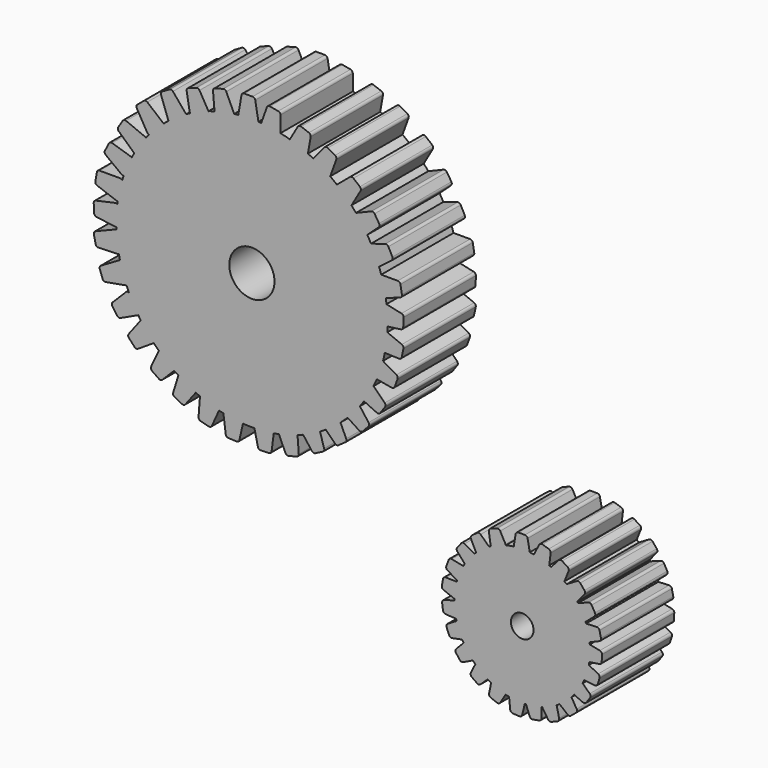
from build123d import *

# Parameters (mm, degrees)
F0_R     = 6.35
F1_DEPTH = 12.7
F0_R_2   = 3.175
F2_DEPTH = 25.4


# Not quite as in the source:
# - a feature names something its author has since deleted; it is built from what else it names


with BuildPart() as f1:
    # F0 (on Front) → F1 (new body)
    with BuildSketch(Plane.XZ):
        with BuildLine():
            Line((-1.757472486, 40.9747326897), (-0.3893329932, 41.4726947414))
            ThreePointArc((-0.3893329932, 41.4726947414), (-0.9286789103, 44.1840079153), (-1.6632014652, 46.8490763501))
            Line((-1.6632014652, 46.8490763501), (-2.7932777673, 46.8490763501))
            ThreePointArc((-2.7932777673, 46.8490763501), (-3.3770036329, 46.5768805087), (-3.5437012751, 45.9547564387))
            Line((-3.5437012751, 45.9547564387), (-2.768515343, 41.5584585553))
            ThreePointArc((-2.768515343, 41.5584585553), (-2.3990918352, 41.030867109), (-1.757472486, 40.9747326897))
        make_face()
        with BuildLine():
            Line((-24.8343352323, -5.0800769341), (-25.1807019478, -0.4779456677))
            ThreePointArc((-25.1807019478, -0.4779456677), (-27.7757681046, -1.3020204716), (-30.4230615323, -1.9386562762))
            Line((-30.4230615323, -1.9386562762), (-28.5737988695, -6.0335388506))
            ThreePointArc((-28.5737988695, -6.0335388506), (-28.2097311384, -6.4065595844), (-27.6910659701, -6.458291818))
            Line((-27.6910659701, -6.458291818), (-25.4059202071, -5.8756415586))
            ThreePointArc((-25.4059202071, -5.8756415586), (-24.9753467984, -5.5818792049), (-24.8343352323, -5.0800769341))
        make_face()
        with BuildLine():
            ThreePointArc((0.0896368674, 34.6132318585), (0.0957281106, 35.006533234), (0.0977585971, 35.3998765349))
            ThreePointArc((0.0977585971, 35.3998765349), (0.0271905358, 37.7177001734), (-0.1842522385, 40.0269377582))
            Line((-0.1842522385, 40.0269377582), (-1.40801912, 40.2964548052))
            ThreePointArc((-1.40801912, 40.2964548052), (-2.0366277798, 40.156177882), (-2.3332312801, 39.5844674432))
            Line((-2.3332312801, 39.5844674432), (-2.5198951773, 35.1681897237))
            ThreePointArc((-2.5198951773, 35.1681897237), (-2.2725926276, 34.573489874), (-1.6580630976, 34.3806689231))
            Line((-1.6580630976, 34.3806689231), (0.0896368674, 34.6132318585))
        make_face()
        with BuildLine():
            ThreePointArc((-76.0691807286, 33.8130147361), (-75.8300529447, 30.8538151675), (-75.361238122, 27.922218871))
            Line((-75.361238122, 27.922218871), (-75.1012664563, 27.9322852077))
            ThreePointArc((-75.1012664563, 27.9322852077), (-74.5285094671, 28.2268626911), (-74.3860078154, 28.8549707563))
            Line((-74.3860078154, 28.8549707563), (-75.3294811586, 33.2122875626))
            ThreePointArc((-75.3294811586, 33.2122875626), (-75.5938457194, 33.6425393555), (-76.0691807286, 33.8130147361))
        make_face()
        with BuildLine():
            Line((-3.1541498724, 47.9642560193), (-2.2736241306, 48.6315018249))
            ThreePointArc((-2.2736241306, 48.6315018249), (-3.3108628149, 51.1516463297), (-4.5255958714, 53.5911987508))
            Line((-4.5255958714, 53.5911987508), (-5.8332779518, 53.1875496492))
            ThreePointArc((-5.8332779518, 53.1875496492), (-6.3107540994, 52.7552962619), (-6.2865445456, 52.1116811907))
            Line((-6.2865445456, 52.1116811907), (-4.2923823896, 48.2238138779))
            ThreePointArc((-4.2923823896, 48.2238138779), (-3.7837830396, 47.8286516788), (-3.1541498724, 47.9642560193))
        make_face()
        with BuildLine():
            Line((-17.6963946169, -1.3683205653), (-18.8767527981, 2.4480073068))
            ThreePointArc((-18.8767527981, 2.4480073068), (-21.1986845934, 1.2055717672), (-23.6008947628, 0.1264982596))
            Line((-23.6008947628, 0.1264982596), (-21.1291628676, -3.1314938572))
            ThreePointArc((-21.1291628676, -3.1314938572), (-20.6910940628, -3.4139571344), (-20.1739499944, -3.3487513584))
            Line((-20.1739499944, -3.3487513584), (-18.0762224632, -2.2712952395))
            ThreePointArc((-18.0762224632, -2.2712952395), (-17.7219805882, -1.8889309175), (-17.6963946169, -1.3683205653))
        make_face()
        with BuildLine():
            ThreePointArc((-75.0611048511, 26.553937358), (-74.2600521977, 23.6959816119), (-73.2389565027, 20.9090549925))
            ThreePointArc((-73.2389565027, 20.9090549925), (-72.7173326069, 21.2826770925), (-72.6659881309, 21.9222462498))
            Line((-72.6659881309, 21.9222462498), (-74.2011624613, 26.0703961395))
            ThreePointArc((-74.2011624613, 26.0703961395), (-74.5423174876, 26.4701197534), (-75.0611048511, 26.553937358))
        make_face()
        with BuildLine():
            Line((-6.5940966355, 54.4887193588), (-5.5842373836, 55.4169446372))
            ThreePointArc((-5.5842373836, 55.4169446372), (-7.0921899631, 57.6749460071), (-8.757129668, 59.8198159209))
            Line((-8.757129668, 59.8198159209), (-9.7404233247, 59.4107504158))
            ThreePointArc((-9.7404233247, 59.4107504158), (-10.1748204192, 58.9352237324), (-10.0897709159, 58.2967935919))
            Line((-10.0897709159, 58.2967935919), (-7.7517935247, 54.6393230026))
            ThreePointArc((-7.7517935247, 54.6393230026), (-7.2080588963, 54.2940997181), (-6.5940966355, 54.4887193588))
        make_face()
        with BuildLine():
            Line((-11.4894055802, 3.0583391146), (-13.117311746, 6.549395153))
            ThreePointArc((-13.117311746, 6.549395153), (-15.1319475431, 4.9275996464), (-17.2519690113, 3.4462195349))
            Line((-17.2519690113, 3.4462195349), (-14.6505978994, 0.844848423))
            ThreePointArc((-14.6505978994, 0.844848423), (-14.1781952081, 0.6245634304), (-13.6747172876, 0.7594699326))
            Line((-13.6747172876, 0.7594699326), (-11.7429468695, 2.1121101414))
            ThreePointArc((-11.7429468695, 2.1121101414), (-11.4439766343, 2.5390838868), (-11.4894055802, 3.0583391146))
        make_face()
        with BuildLine():
            Line((2.6020832503, 23.4633030424), (-1.166559288, 25.6662994365))
            ThreePointArc((-1.166559288, 25.6662994365), (-1.9412722958, 23.1028644157), (-2.8941370725, 20.6001802432))
            Line((-2.8941370725, 20.6001802432), (1.2626647425, 19.8440992652))
            ThreePointArc((1.2626647425, 19.8440992652), (1.7764650698, 19.9318432361), (2.1136582181, 20.3293235016))
            Line((2.1136582181, 20.3293235016), (2.932162374, 22.5409797655))
            ThreePointArc((2.932162374, 22.5409797655), (2.9349719218, 23.062210892), (2.6020832503, 23.4633030424))
        make_face()
        with BuildLine():
            ThreePointArc((-58.6634660467, 3.3885692168), (-56.2704157813, 1.9651071342), (-53.7797966455, 0.7202175031))
            Line((-53.7797966455, 0.7202175031), (-53.4749955725, 1.1219760817))
            ThreePointArc((-53.4749955725, 1.1219760817), (-53.3390369996, 1.7515328534), (-53.7339129801, 2.2603544551))
            Line((-53.7339129801, 2.2603544551), (-57.4810229109, 4.1849831131))
            ThreePointArc((-57.4810229109, 4.1849831131), (-58.124624259, 4.2095547836), (-58.5571462229, 3.7323219126))
            Line((-58.5571462229, 3.7323219126), (-58.6634660467, 3.3885692168))
        make_face()
        with BuildLine():
            Line((-22.4147191758, 69.2607800844), (-22.2669644065, 70.0987390213))
            ThreePointArc((-22.2669644065, 70.0987390213), (-24.7714102718, 71.1287879035), (-27.3426957081, 71.9783413138))
            Line((-27.3426957081, 71.9783413138), (-27.7834949358, 71.2148546555))
            ThreePointArc((-27.7834949358, 71.2148546555), (-27.8396293552, 70.5732353062), (-27.3842029274, 70.1178088784))
            Line((-27.3842029274, 70.1178088784), (-23.4257620329, 68.6770542187))
            ThreePointArc((-23.4257620329, 68.6770542187), (-22.7841426836, 68.7331886381), (-22.4147191758, 69.2607800844))
        make_face()
        with BuildLine():
            Line((-10.3777093051, 60.6783340478), (-10.0344464864, 61.2728826902))
            ThreePointArc((-10.0344464864, 61.2728826902), (-12.0065419943, 63.2536664433), (-14.1185481463, 65.0845391813))
            Line((-14.1185481463, 65.0845391813), (-14.8736841245, 64.4509048605))
            ThreePointArc((-14.8736841245, 64.4509048605), (-15.1458799659, 63.8671789948), (-14.8736841245, 63.2834531292))
            Line((-14.8736841245, 63.2834531292), (-11.5274248214, 60.4756081821))
            ThreePointArc((-11.5274248214, 60.4756081821), (-10.9053007514, 60.30891054), (-10.3777093051, 60.6783340478))
        make_face()
        with BuildLine():
            Line((-5.207969894, 9.1186594653), (-7.6623129761, 12.3542968491))
            ThreePointArc((-7.6623129761, 12.3542968491), (-9.320562803, 10.3205760523), (-11.1148661628, 8.4058206578))
            Line((-11.1148661628, 8.4058206578), (-7.830914341, 6.2879633764))
            ThreePointArc((-7.830914341, 6.2879633764), (-7.3226659177, 6.172320301), (-6.8589911012, 6.4104283549))
            Line((-6.8589911012, 6.4104283549), (-5.2561381332, 8.1402361031))
            ThreePointArc((-5.2561381332, 8.1402361031), (-5.0539955234, 8.6206818816), (-5.207969894, 9.1186594653))
        make_face()
        with BuildLine():
            ThreePointArc((-64.1725706464, 7.7100974226), (-62.0727974784, 5.8665338488), (-59.8435560221, 4.1818212511))
            Line((-59.8435560221, 4.1818212511), (-59.4052585956, 4.6201186776))
            ThreePointArc((-59.4052585956, 4.6201186776), (-59.1849736029, 5.2253467209), (-59.5070087183, 5.7831279026))
            Line((-59.5070087183, 5.7831279026), (-62.9576742649, 8.1993099302))
            ThreePointArc((-62.9576742649, 8.1993099302), (-63.5919596218, 8.3111515521), (-64.0853460431, 7.8971511879))
            Line((-64.0853460431, 7.8971511879), (-64.1725706464, 7.7100974226))
        make_face()
        with BuildLine():
            Line((-16.3259688987, 65.6350036516), (-16.0074897376, 66.5100179551))
            ThreePointArc((-16.0074897376, 66.5100179551), (-18.3466451023, 68.0383129875), (-20.7915160489, 69.3910655814))
            Line((-20.7915160489, 69.3910655814), (-21.457320418, 68.5975908326))
            ThreePointArc((-21.457320418, 68.5975908326), (-21.6240180601, 67.9754667626), (-21.2545945523, 67.4478753163))
            Line((-21.2545945523, 67.4478753163), (-17.4230146757, 65.2357116431))
            ThreePointArc((-17.4230146757, 65.2357116431), (-16.7813953265, 65.1795772238), (-16.3259688987, 65.6350036516))
        make_face()
        with BuildLine():
            Line((-0.6777773465, 15.4575499219), (-3.8107741652, 18.5905467406))
            ThreePointArc((-3.8107741652, 18.5905467406), (-5.0722603995, 16.2367256688), (-6.4955330194, 13.9770539656))
            Line((-6.4955330194, 13.9770539656), (-2.8912680381, 12.2963576028))
            ThreePointArc((-2.8912680381, 12.2963576028), (-2.3720128103, 12.2509286569), (-1.9450390649, 12.549898892))
            Line((-1.9450390649, 12.549898892), (-0.5923988561, 14.4816693102))
            ThreePointArc((-0.5923988561, 14.4816693102), (-0.4574923539, 14.9851472306), (-0.6777773465, 15.4575499219))
        make_face()
        with BuildLine():
            ThreePointArc((-76.0884323262, 34.3741763108), (-76.0561217743, 37.2739599584), (-75.8033490381, 40.1628862501))
            ThreePointArc((-75.8033490381, 40.1628862501), (-76.0986776972, 40.2971855357), (-76.4231076296, 40.2964548052))
            Line((-76.4231076296, 40.2964548052), (-81.8571995919, 39.0996742413))
            ThreePointArc((-81.8571995919, 39.0996742413), (-82.2971970273, 38.8202247152), (-82.4546279247, 38.3233290589))
            Line((-82.4546279247, 38.3233290589), (-82.3495712429, 35.8377949505))
            ThreePointArc((-82.3495712429, 35.8377949505), (-82.1507719359, 35.3559561639), (-81.6887628296, 35.1146319703))
            Line((-81.6887628296, 35.1146319703), (-76.1730636519, 34.3806689231))
            ThreePointArc((-76.1730636519, 34.3806689231), (-76.1308384617, 34.3762433048), (-76.0884323262, 34.3741763108))
        make_face()
        with BuildLine():
            Line((-29.9811336016, 71.8112511766), (-29.9811336016, 72.645974715))
            ThreePointArc((-29.9811336016, 72.645974715), (-32.6702976431, 73.1249395003), (-35.3868669024, 73.4100043461))
            Line((-35.3868669024, 73.4100043461), (-35.6076670825, 72.8033608372))
            ThreePointArc((-35.6076670825, 72.8033608372), (-35.5515326632, 72.161741488), (-35.0239412169, 71.7923179802))
            Line((-35.0239412169, 71.7923179802), (-30.875453513, 71.0608276688))
            ThreePointArc((-30.875453513, 71.0608276688), (-30.253329443, 71.227525311), (-29.9811336016, 71.8112511766))
        make_face()
        with BuildLine():
            Line((4.1290907018, 31.4700232345), (0.0309104009, 33.1439146842))
            ThreePointArc((0.0309104009, 33.1439146842), (-0.2204609236, 30.4859103346), (-0.6573608201, 27.8520361643))
            Line((-0.6573608201, 27.8520361643), (3.3124186443, 27.6983227333))
            ThreePointArc((3.3124186443, 27.6983227333), (3.8087537974, 27.857511918), (4.0866437478, 28.298495995))
            Line((4.0866437478, 28.298495995), (4.5857032047, 30.6033413567))
            ThreePointArc((4.5857032047, 30.6033413567), (4.5151201563, 31.1197789754), (4.1290907018, 31.4700232345))
        make_face()
        with BuildLine():
            Line((-81.1435453938, 27.6983227333), (-75.361238122, 27.922218871))
            ThreePointArc((-75.361238122, 27.922218871), (-75.8300529447, 30.8538151675), (-76.0691807286, 33.8130147361))
            ThreePointArc((-76.0691807286, 33.8130147361), (-76.2185638148, 33.7992357617), (-76.3623524, 33.7564571535))
            Line((-76.3623524, 33.7564571535), (-81.9602174513, 31.4700232345))
            ThreePointArc((-81.9602174513, 31.4700232345), (-82.3462469058, 31.1197789754), (-82.4168299543, 30.6033413567))
            Line((-82.4168299543, 30.6033413567), (-81.9177704974, 28.298495995))
            ThreePointArc((-81.9177704974, 28.298495995), (-81.6398805469, 27.857511918), (-81.1435453938, 27.6983227333))
        make_face()
        with BuildLine():
            ThreePointArc((-46.0190922885, -1.8471381357), (-43.2862430647, -2.3319313523), (-40.52535239, -2.6164871911))
            Line((-40.52535239, -2.6164871911), (-40.3481192857, -1.8195910708))
            ThreePointArc((-40.3481192857, -1.8195910708), (-40.4870963261, -1.1906937465), (-41.0581923463, -0.8929089281))
            Line((-41.0581923463, -0.8929089281), (-45.2665425837, -0.7063169032))
            ThreePointArc((-45.2665425837, -0.7063169032), (-45.8617524348, -0.9523894444), (-46.0558434495, -1.5665190238))
            Line((-46.0558434495, -1.5665190238), (-46.0190922885, -1.8471381357))
        make_face()
        with BuildLine():
            ThreePointArc((-41.8303742214, 73.3070710912), (-39.0040716767, 73.4867028152), (-36.172233945, 73.4559019804))
            Line((-36.172233945, 73.4559019804), (-37.0634814029, 78.5104174853))
            ThreePointArc((-37.0634814029, 78.5104174853), (-37.3241007521, 78.9618234396), (-37.8139049107, 79.1400975739))
            Line((-37.8139049107, 79.1400975739), (-40.1721611485, 79.1400975739))
            ThreePointArc((-40.1721611485, 79.1400975739), (-40.6619653071, 78.9618234396), (-40.9225846563, 78.5104174853))
            Line((-40.9225846563, 78.5104174853), (-41.818895476, 73.4271862288))
            ThreePointArc((-41.818895476, 73.4271862288), (-41.8270161089, 73.367356224), (-41.8303742214, 73.3070710912))
        make_face()
        with BuildLine():
            ThreePointArc((-0.1842522385, 40.0269377582), (0.0271905358, 37.7177001734), (0.0977585971, 35.3998765349))
            ThreePointArc((0.0977585971, 35.3998765349), (0.0957281106, 35.006533234), (0.0896368674, 34.6132318585))
            Line((0.0896368674, 34.6132318585), (3.8576360801, 35.1146319703))
            ThreePointArc((3.8576360801, 35.1146319703), (4.3196451864, 35.3559561639), (4.5184444934, 35.8377949505))
            Line((4.5184444934, 35.8377949505), (4.6235011752, 38.3233290589))
            ThreePointArc((4.6235011752, 38.3233290589), (4.4660702778, 38.8202247152), (4.0260728424, 39.0996742413))
            Line((4.0260728424, 39.0996742413), (-0.1842522385, 40.0269377582))
        make_face()
        with BuildLine():
            ThreePointArc((-73.2442558578, 20.908071718), (-73.2416053109, 20.9085586698), (-73.2389565027, 20.9090549925))
            ThreePointArc((-73.2389565027, 20.9090549925), (-74.2600521977, 23.6959816119), (-75.0611048511, 26.553937358))
            ThreePointArc((-75.0611048511, 26.553937358), (-75.1845333609, 26.518958615), (-75.3003445401, 26.4637691211))
            Line((-75.3003445401, 26.4637691211), (-80.4332099998, 23.4633030424))
            ThreePointArc((-80.4332099998, 23.4633030424), (-80.7660986713, 23.062210892), (-80.7632891235, 22.5409797655))
            Line((-80.7632891235, 22.5409797655), (-79.9447849676, 20.3293235016))
            ThreePointArc((-79.9447849676, 20.3293235016), (-79.6075918193, 19.9318432361), (-79.0937914921, 19.8440992652))
            Line((-79.0937914921, 19.8440992652), (-73.2442558578, 20.908071718))
        make_face()
        with BuildLine():
            ThreePointArc((-37.2886596196, -2.6934404779), (-34.56474029, -2.5447355477), (-31.8584437149, -2.2015030936))
            Line((-31.8584437149, -2.2015030936), (-31.7752833001, -1.5665190238))
            ThreePointArc((-31.7752833001, -1.5665190238), (-31.9693743147, -0.9523894444), (-32.5645841658, -0.7063169032))
            Line((-32.5645841658, -0.7063169032), (-36.7729344032, -0.8929089281))
            ThreePointArc((-36.7729344032, -0.8929089281), (-37.3440304234, -1.1906937465), (-37.4830074638, -1.8195910708))
            Line((-37.4830074638, -1.8195910708), (-37.2886596196, -2.6934404779))
        make_face()
        with BuildLine():
            ThreePointArc((-43.5182135727, 72.2138066545), (-43.0490250068, 72.5803242408), (-42.986667335, 73.1724260667))
            ThreePointArc((-42.986667335, 73.1724260667), (-45.7659870186, 72.7004697476), (-48.5028012864, 72.0242979247))
            Line((-48.5028012864, 72.0242979247), (-48.4839741884, 71.8091032096))
            ThreePointArc((-48.4839741884, 71.8091032096), (-48.1619390729, 71.2513220279), (-47.5276537161, 71.139480406))
            Line((-47.5276537161, 71.139480406), (-43.5182135727, 72.2138066545))
        make_face()
        with BuildLine():
            ThreePointArc((-70.1010466381, 14.5527327289), (-70.0240696264, 14.5941603025), (-69.9523439091, 14.6441315509))
            ThreePointArc((-69.9523439091, 14.6441315509), (-71.3543573298, 16.9812348045), (-72.5857124564, 19.412583772))
            ThreePointArc((-72.5857124564, 19.412583772), (-73.0078539085, 19.4371207954), (-73.3780791484, 19.2328201765))
            Line((-73.3780791484, 19.2328201765), (-77.153349403, 15.4575499219))
            ThreePointArc((-77.153349403, 15.4575499219), (-77.3736343957, 14.9851472306), (-77.2387278935, 14.4816693102))
            Line((-77.2387278935, 14.4816693102), (-75.8860876846, 12.549898892))
            ThreePointArc((-75.8860876846, 12.549898892), (-75.4591139392, 12.2509286569), (-74.9398587114, 12.2963576028))
            Line((-74.9398587114, 12.2963576028), (-70.1010466381, 14.5527327289))
        make_face()
        with BuildLine():
            ThreePointArc((-30.4230615323, -1.9386562762), (-27.7757681046, -1.3020204716), (-25.1807019478, -0.4779456677))
            Line((-25.1807019478, -0.4779456677), (-25.2350299841, 0.2439041615))
            ThreePointArc((-25.2350299841, 0.2439041615), (-25.550266789, 0.8055554939), (-26.1831469834, 0.9250926087))
            Line((-26.1831469834, 0.9250926087), (-30.2650366734, -0.1156786741))
            ThreePointArc((-30.2650366734, -0.1156786741), (-30.7634149634, -0.5236560539), (-30.7712375483, -1.1676787783))
            Line((-30.7712375483, -1.1676787783), (-30.4230615323, -1.9386562762))
        make_face()
        with BuildLine():
            Line((-70.0002124085, 6.2879633764), (-65.5959796557, 9.1283023675))
            ThreePointArc((-65.5959796557, 9.1283023675), (-67.4866835263, 11.2694461064), (-69.2116602667, 13.546222969))
            ThreePointArc((-69.2116602667, 13.546222969), (-69.31139016, 13.4670625555), (-69.3965465211, 13.3724009643))
            Line((-69.3965465211, 13.3724009643), (-72.6231568555, 9.1186594653))
            ThreePointArc((-72.6231568555, 9.1186594653), (-72.7771312261, 8.6206818816), (-72.5749886163, 8.1402361031))
            Line((-72.5749886163, 8.1402361031), (-70.9721356483, 6.4104283549))
            ThreePointArc((-70.9721356483, 6.4104283549), (-70.5084608318, 6.172320301), (-70.0002124085, 6.2879633764))
        make_face()
        with BuildLine():
            ThreePointArc((-23.6008947628, 0.1264982596), (-21.1986845934, 1.2055717672), (-18.8767527981, 2.4480073068))
            Line((-18.8767527981, 2.4480073068), (-19.2739805266, 3.7323219126))
            ThreePointArc((-19.2739805266, 3.7323219126), (-19.7065024905, 4.2095547836), (-20.3501038386, 4.1849831131))
            Line((-20.3501038386, 4.1849831131), (-24.0972137694, 2.2603544551))
            ThreePointArc((-24.0972137694, 2.2603544551), (-24.4920897499, 1.7515328534), (-24.356131177, 1.1219760817))
            Line((-24.356131177, 1.1219760817), (-23.6008947628, 0.1264982596))
        make_face()
        with BuildLine():
            Line((-63.1805288502, 0.844848423), (-59.8435560221, 4.1818212511))
            ThreePointArc((-59.8435560221, 4.1818212511), (-62.0727974784, 5.8665338488), (-64.1725706464, 7.7100974226))
            Line((-64.1725706464, 7.7100974226), (-66.3417211693, 3.0583391146))
            ThreePointArc((-66.3417211693, 3.0583391146), (-66.3871501152, 2.5390838868), (-66.0881798801, 2.1121101414))
            Line((-66.0881798801, 2.1121101414), (-64.1564094619, 0.7594699326))
            ThreePointArc((-64.1564094619, 0.7594699326), (-63.6529315414, 0.6245634304), (-63.1805288502, 0.844848423))
        make_face()
        with BuildLine():
            ThreePointArc((-17.2519690113, 3.4462195349), (-15.1319475431, 4.9275996464), (-13.117311746, 6.549395153))
            Line((-13.117311746, 6.549395153), (-13.7457807064, 7.8971511879))
            ThreePointArc((-13.7457807064, 7.8971511879), (-14.2391671277, 8.3111515521), (-14.8734524846, 8.1993099302))
            Line((-14.8734524846, 8.1993099302), (-18.3241180312, 5.7831279026))
            ThreePointArc((-18.3241180312, 5.7831279026), (-18.6461531466, 5.2253467209), (-18.425868154, 4.6201186776))
            Line((-18.425868154, 4.6201186776), (-17.2519690113, 3.4462195349))
        make_face()
        with BuildLine():
            Line((-1.40801912, 40.2964548052), (-0.1842522385, 40.0269377582))
            ThreePointArc((-0.1842522385, 40.0269377582), (-0.2798656755, 40.7507988369), (-0.3893329932, 41.4726947414))
            Line((-0.3893329932, 41.4726947414), (-1.757472486, 40.9747326897))
            ThreePointArc((-1.757472486, 40.9747326897), (-2.3990918352, 41.030867109), (-2.768515343, 41.5584585553))
            Line((-2.768515343, 41.5584585553), (-3.5437012751, 45.9547564387))
            ThreePointArc((-3.5437012751, 45.9547564387), (-3.3770036329, 46.5768805087), (-2.7932777673, 46.8490763501))
            Line((-2.7932777673, 46.8490763501), (-1.6632014652, 46.8490763501))
            ThreePointArc((-1.6632014652, 46.8490763501), (-1.9573934482, 47.7440628558), (-2.2736241306, 48.6315018249))
            Line((-2.2736241306, 48.6315018249), (-3.1541498724, 47.9642560193))
            ThreePointArc((-3.1541498724, 47.9642560193), (-3.7837830396, 47.8286516788), (-4.2923823896, 48.2238138779))
            Line((-4.2923823896, 48.2238138779), (-6.2865445456, 52.1116811907))
            ThreePointArc((-6.2865445456, 52.1116811907), (-6.3107540994, 52.7552962619), (-5.8332779518, 53.1875496492))
            Line((-5.8332779518, 53.1875496492), (-4.5255958714, 53.5911987508))
            ThreePointArc((-4.5255958714, 53.5911987508), (-5.0422725488, 54.5114032437), (-5.5842373836, 55.4169446372))
            Line((-5.5842373836, 55.4169446372), (-6.5940966355, 54.4887193588))
            ThreePointArc((-6.5940966355, 54.4887193588), (-7.2080588963, 54.2940997181), (-7.7517935247, 54.6393230026))
            Line((-7.7517935247, 54.6393230026), (-10.0897709159, 58.2967935919))
            ThreePointArc((-10.0897709159, 58.2967935919), (-10.1748204192, 58.9352237324), (-9.7404233247, 59.4107504158))
            Line((-9.7404233247, 59.4107504158), (-8.757129668, 59.8198159209))
            ThreePointArc((-8.757129668, 59.8198159209), (-9.3865634861, 60.5544581726), (-10.0344464864, 61.2728826902))
            Line((-10.0344464864, 61.2728826902), (-10.3777093051, 60.6783340478))
            ThreePointArc((-10.3777093051, 60.6783340478), (-10.9053007514, 60.30891054), (-11.5274248214, 60.4756081821))
            Line((-11.5274248214, 60.4756081821), (-14.8736841245, 63.2834531292))
            ThreePointArc((-14.8736841245, 63.2834531292), (-15.1458799659, 63.8671789948), (-14.8736841245, 64.4509048605))
            Line((-14.8736841245, 64.4509048605), (-14.1185481463, 65.0845391813))
            ThreePointArc((-14.1185481463, 65.0845391813), (-15.051948931, 65.8119477478), (-16.0074897376, 66.5100179551))
            Line((-16.0074897376, 66.5100179551), (-16.3259688987, 65.6350036516))
            ThreePointArc((-16.3259688987, 65.6350036516), (-16.7813953265, 65.1795772238), (-17.4230146757, 65.2357116431))
            Line((-17.4230146757, 65.2357116431), (-21.2545945523, 67.4478753163))
            ThreePointArc((-21.2545945523, 67.4478753163), (-21.6240180601, 67.9754667626), (-21.457320418, 68.5975908326))
            Line((-21.457320418, 68.5975908326), (-20.7915160489, 69.3910655814))
            ThreePointArc((-20.7915160489, 69.3910655814), (-21.5254404955, 69.7528244704), (-22.2669644065, 70.0987390213))
            Line((-22.2669644065, 70.0987390213), (-22.4147191758, 69.2607800844))
            ThreePointArc((-22.4147191758, 69.2607800844), (-22.7841426836, 68.7331886381), (-23.4257620329, 68.6770542187))
            Line((-23.4257620329, 68.6770542187), (-27.3842029274, 70.1178088784))
            ThreePointArc((-27.3842029274, 70.1178088784), (-27.8396293552, 70.5732353062), (-27.7834949358, 71.2148546555))
            Line((-27.7834949358, 71.2148546555), (-27.3426957081, 71.9783413138))
            ThreePointArc((-27.3426957081, 71.9783413138), (-28.6559513716, 72.3357244696), (-29.9811336016, 72.645974715))
            Line((-29.9811336016, 72.645974715), (-29.9811336016, 71.8112511766))
            ThreePointArc((-29.9811336016, 71.8112511766), (-30.253329443, 71.227525311), (-30.875453513, 71.0608276688))
            Line((-30.875453513, 71.0608276688), (-35.0239412169, 71.7923179802))
            ThreePointArc((-35.0239412169, 71.7923179802), (-35.5515326632, 72.161741488), (-35.6076670825, 72.8033608372))
            Line((-35.6076670825, 72.8033608372), (-35.3868669024, 73.4100043461))
            ThreePointArc((-35.3868669024, 73.4100043461), (-35.779431956, 73.4349802966), (-36.172233945, 73.4559019804))
            Line((-36.172233945, 73.4559019804), (-36.1671705832, 73.4271862288))
            ThreePointArc((-36.1671705832, 73.4271862288), (-36.3338682254, 72.8050621589), (-36.917594091, 72.5328663174))
            Line((-36.917594091, 72.5328663174), (-41.0684719682, 72.5328663174))
            ThreePointArc((-41.0684719682, 72.5328663174), (-41.6115852333, 72.7603834073), (-41.8303742214, 73.3070710912))
            ThreePointArc((-41.8303742214, 73.3070710912), (-42.4090350507, 73.2441650042), (-42.986667335, 73.1724260667))
            ThreePointArc((-42.986667335, 73.1724260667), (-43.0490250068, 72.5803242408), (-43.5182135727, 72.2138066545))
            Line((-43.5182135727, 72.2138066545), (-47.5276537161, 71.139480406))
            ThreePointArc((-47.5276537161, 71.139480406), (-48.1619390729, 71.2513220279), (-48.4839741884, 71.8091032096))
            Line((-48.4839741884, 71.8091032096), (-48.5028012864, 72.0242979247))
            ThreePointArc((-48.5028012864, 72.0242979247), (-49.358330583, 71.7681214546), (-50.2076205138, 71.4919632127))
            Line((-50.2076205138, 71.4919632127), (-50.0476318137, 71.2148546555))
            ThreePointArc((-50.0476318137, 71.2148546555), (-49.9914973943, 70.5732353062), (-50.4469238222, 70.1178088784))
            Line((-50.4469238222, 70.1178088784), (-54.4053647167, 68.6770542187))
            ThreePointArc((-54.4053647167, 68.6770542187), (-55.0469840659, 68.7331886381), (-55.4164075737, 69.2607800844))
            Line((-55.4164075737, 69.2607800844), (-55.4206936268, 69.2850874996))
            ThreePointArc((-55.4206936268, 69.2850874996), (-55.9511697125, 69.007107491), (-56.4772108043, 68.7208234845))
            Line((-56.4772108043, 68.7208234845), (-56.3738063316, 68.5975908326))
            ThreePointArc((-56.3738063316, 68.5975908326), (-56.2071086894, 67.9754667626), (-56.5765321972, 67.4478753163))
            Line((-56.5765321972, 67.4478753163), (-60.4081120738, 65.2357116431))
            ThreePointArc((-60.4081120738, 65.2357116431), (-60.9540887127, 65.1516964529), (-61.4133642691, 65.4586410828))
            ThreePointArc((-61.4133642691, 65.4586410828), (-62.1253885837, 64.8902778563), (-62.8236195355, 64.3050523274))
            ThreePointArc((-62.8236195355, 64.3050523274), (-62.6917015468, 63.7682073061), (-62.957442625, 63.2834531292))
            Line((-62.957442625, 63.2834531292), (-66.3037019281, 60.4756081821))
            ThreePointArc((-66.3037019281, 60.4756081821), (-66.5551734404, 60.3355650586), (-66.8406517783, 60.2987939214))
            ThreePointArc((-66.8406517783, 60.2987939214), (-67.314748998, 59.7388760724), (-67.7779767525, 59.1699330008))
            ThreePointArc((-67.7779767525, 59.1699330008), (-67.6220593446, 58.7391347606), (-67.7413558336, 58.2967935919))
            Line((-67.7413558336, 58.2967935919), (-70.0793332248, 54.6393230026))
            ThreePointArc((-70.0793332248, 54.6393230026), (-70.5114739264, 54.3172105271), (-71.048626444, 54.3615862604))
            ThreePointArc((-71.048626444, 54.3615862604), (-71.4104399128, 53.7165976477), (-71.7596662621, 53.0647078921))
            ThreePointArc((-71.7596662621, 53.0647078921), (-71.4792905177, 52.6272005596), (-71.5445822039, 52.1116811907))
            Line((-71.5445822039, 52.1116811907), (-73.53874436, 48.2238138779))
            ThreePointArc((-73.53874436, 48.2238138779), (-73.7362773682, 47.9801562359), (-74.0152263502, 47.8367135599))
            ThreePointArc((-74.0152263502, 47.8367135599), (-74.2301685861, 47.1959475761), (-74.433710903, 46.5514696975))
            ThreePointArc((-74.433710903, 46.5514696975), (-74.2977638847, 46.2685096667), (-74.2874254745, 45.9547564387))
            Line((-74.2874254745, 45.9547564387), (-75.0626114065, 41.5584585553))
            ThreePointArc((-75.0626114065, 41.5584585553), (-75.2803227059, 41.1459283011), (-75.6976523835, 40.9375647709))
            ThreePointArc((-75.6976523835, 40.9375647709), (-75.752487925, 40.5504966448), (-75.8033490381, 40.1628862501))
            ThreePointArc((-75.8033490381, 40.1628862501), (-75.585399657, 39.9081198397), (-75.4978954694, 39.5844674432))
            Line((-75.4978954694, 39.5844674432), (-75.3112315722, 35.1681897237))
            ThreePointArc((-75.3112315722, 35.1681897237), (-75.5280020725, 34.6029915137), (-76.0884323262, 34.3741763108))
            ThreePointArc((-76.0884323262, 34.3741763108), (-76.0798402933, 34.0935600583), (-76.0691807286, 33.8130147361))
            ThreePointArc((-76.0691807286, 33.8130147361), (-75.5938457194, 33.6425393555), (-75.3294811586, 33.2122875626))
            Line((-75.3294811586, 33.2122875626), (-74.3860078154, 28.8549707563))
            ThreePointArc((-74.3860078154, 28.8549707563), (-74.5285094671, 28.2268626911), (-75.1012664563, 27.9322852077))
            Line((-75.1012664563, 27.9322852077), (-75.361238122, 27.922218871))
            ThreePointArc((-75.361238122, 27.922218871), (-75.2174604208, 27.2366986335), (-75.0611048511, 26.553937358))
            ThreePointArc((-75.0611048511, 26.553937358), (-74.5423174876, 26.4701197534), (-74.2011624613, 26.0703961395))
            Line((-74.2011624613, 26.0703961395), (-72.6659881309, 21.9222462498))
            ThreePointArc((-72.6659881309, 21.9222462498), (-72.7173326069, 21.2826770925), (-73.2389565027, 20.9090549925))
            ThreePointArc((-73.2389565027, 20.9090549925), (-72.9203521071, 20.1573195038), (-72.5857124564, 19.412583772))
            ThreePointArc((-72.5857124564, 19.412583772), (-72.3783715543, 19.300818088), (-72.2150699234, 19.1310700538))
            Line((-72.2150699234, 19.1310700538), (-69.7988878958, 15.6804045072))
            ThreePointArc((-69.7988878958, 15.6804045072), (-69.669301767, 15.1317160934), (-69.9523439091, 14.6441315509))
            ThreePointArc((-69.9523439091, 14.6441315509), (-69.5867729925, 14.0919586577), (-69.2116602667, 13.546222969))
            ThreePointArc((-69.2116602667, 13.546222969), (-68.699658422, 13.6685836287), (-68.230506964, 13.4298056364))
            Line((-68.230506964, 13.4298056364), (-65.3673771319, 10.3399001575))
            ThreePointArc((-65.3673771319, 10.3399001575), (-65.1702907197, 9.7267252978), (-65.5133252099, 9.1816071447))
            Line((-65.5133252099, 9.1816071447), (-65.5959796557, 9.1283023675))
            ThreePointArc((-65.5959796557, 9.1283023675), (-64.8936259852, 8.4098147483), (-64.1725706464, 7.7100974226))
            Line((-64.1725706464, 7.7100974226), (-64.0853460431, 7.8971511879))
            ThreePointArc((-64.0853460431, 7.8971511879), (-63.5919596218, 8.3111515521), (-62.9576742649, 8.1993099302))
            Line((-62.9576742649, 8.1993099302), (-59.5070087183, 5.7831279026))
            ThreePointArc((-59.5070087183, 5.7831279026), (-59.1849736029, 5.2253467209), (-59.4052585956, 4.6201186776))
            Line((-59.4052585956, 4.6201186776), (-59.8435560221, 4.1818212511))
            ThreePointArc((-59.8435560221, 4.1818212511), (-59.2572119544, 3.7796895201), (-58.6634660467, 3.3885692168))
            Line((-58.6634660467, 3.3885692168), (-58.5571462229, 3.7323219126))
            ThreePointArc((-58.5571462229, 3.7323219126), (-58.124624259, 4.2095547836), (-57.4810229109, 4.1849831131))
            Line((-57.4810229109, 4.1849831131), (-53.7339129801, 2.2603544551))
            ThreePointArc((-53.7339129801, 2.2603544551), (-53.3390369996, 1.7515328534), (-53.4749955725, 1.1219760817))
            Line((-53.4749955725, 1.1219760817), (-53.7797966455, 0.7202175031))
            ThreePointArc((-53.7797966455, 0.7202175031), (-53.1915093801, 0.458552314), (-52.5988843658, 0.2068656633))
            Line((-52.5988843658, 0.2068656633), (-52.5960967654, 0.2439041615))
            ThreePointArc((-52.5960967654, 0.2439041615), (-52.2808599606, 0.8055554939), (-51.6479797661, 0.9250926087))
            Line((-51.6479797661, 0.9250926087), (-47.5660900761, -0.1156786741))
            ThreePointArc((-47.5660900761, -0.1156786741), (-47.0677117862, -0.5236560539), (-47.0598892012, -1.1676787783))
            Line((-47.0598892012, -1.1676787783), (-47.2386855108, -1.563593273))
            ThreePointArc((-47.2386855108, -1.563593273), (-46.6300537824, -1.7103761393), (-46.0190922885, -1.8471381357))
            Line((-46.0190922885, -1.8471381357), (-46.0558434495, -1.5665190238))
            ThreePointArc((-46.0558434495, -1.5665190238), (-45.8617524348, -0.9523894444), (-45.2665425837, -0.7063169032))
            Line((-45.2665425837, -0.7063169032), (-41.0581923463, -0.8929089281))
            ThreePointArc((-41.0581923463, -0.8929089281), (-40.4870963261, -1.1906937465), (-40.3481192857, -1.8195910708))
            Line((-40.3481192857, -1.8195910708), (-40.52535239, -2.6164871911))
            ThreePointArc((-40.52535239, -2.6164871911), (-38.9078237773, -2.6893597473), (-37.2886596196, -2.6934404779))
            Line((-37.2886596196, -2.6934404779), (-37.4830074638, -1.8195910708))
            ThreePointArc((-37.4830074638, -1.8195910708), (-37.3440304234, -1.1906937465), (-36.7729344032, -0.8929089281))
            Line((-36.7729344032, -0.8929089281), (-32.5645841658, -0.7063169032))
            ThreePointArc((-32.5645841658, -0.7063169032), (-31.9693743147, -0.9523894444), (-31.7752833001, -1.5665190238))
            Line((-31.7752833001, -1.5665190238), (-31.8584437149, -2.2015030936))
            ThreePointArc((-31.8584437149, -2.2015030936), (-31.1394941119, -2.0769523013), (-30.4230615323, -1.9386562762))
            Line((-30.4230615323, -1.9386562762), (-30.7712375483, -1.1676787783))
            ThreePointArc((-30.7712375483, -1.1676787783), (-30.7634149634, -0.5236560539), (-30.2650366734, -0.1156786741))
            Line((-30.2650366734, -0.1156786741), (-26.1831469834, 0.9250926087))
            ThreePointArc((-26.1831469834, 0.9250926087), (-25.550266789, 0.8055554939), (-25.2350299841, 0.2439041615))
            Line((-25.2350299841, 0.2439041615), (-25.1807019478, -0.4779456677))
            ThreePointArc((-25.1807019478, -0.4779456677), (-24.3874435729, -0.184491944), (-23.6008947628, 0.1264982596))
            Line((-23.6008947628, 0.1264982596), (-24.356131177, 1.1219760817))
            ThreePointArc((-24.356131177, 1.1219760817), (-24.4920897499, 1.7515328534), (-24.0972137694, 2.2603544551))
            Line((-24.0972137694, 2.2603544551), (-20.3501038386, 4.1849831131))
            ThreePointArc((-20.3501038386, 4.1849831131), (-19.7065024905, 4.2095547836), (-19.2739805266, 3.7323219126))
            Line((-19.2739805266, 3.7323219126), (-18.8767527981, 2.4480073068))
            ThreePointArc((-18.8767527981, 2.4480073068), (-18.0581148069, 2.9369466868), (-17.2519690113, 3.4462195349))
            Line((-17.2519690113, 3.4462195349), (-18.425868154, 4.6201186776))
            ThreePointArc((-18.425868154, 4.6201186776), (-18.6461531466, 5.2253467209), (-18.3241180312, 5.7831279026))
            Line((-18.3241180312, 5.7831279026), (-14.8734524846, 8.1993099302))
            ThreePointArc((-14.8734524846, 8.1993099302), (-14.2391671277, 8.3111515521), (-13.7457807064, 7.8971511879))
            Line((-13.7457807064, 7.8971511879), (-13.117311746, 6.549395153))
            ThreePointArc((-13.117311746, 6.549395153), (-12.0994526051, 7.4596629978), (-11.1148661628, 8.4058206578))
            Line((-11.1148661628, 8.4058206578), (-12.3178015396, 9.1816071447))
            ThreePointArc((-12.3178015396, 9.1816071447), (-12.6608360298, 9.7267252978), (-12.4637496177, 10.3399001575))
            Line((-12.4637496177, 10.3399001575), (-9.6006197855, 13.4298056364))
            ThreePointArc((-9.6006197855, 13.4298056364), (-9.0042158879, 13.6729698879), (-8.4345802285, 13.3724009643))
            Line((-8.4345802285, 13.3724009643), (-7.6623129761, 12.3542968491))
            ThreePointArc((-7.6623129761, 12.3542968491), (-7.0682801895, 13.1580231128), (-6.4955330194, 13.9770539656))
            Line((-6.4955330194, 13.9770539656), (-7.7300801114, 14.5527327289))
            ThreePointArc((-7.7300801114, 14.5527327289), (-8.1440804756, 15.0461191503), (-8.0322388537, 15.6804045072))
            Line((-8.0322388537, 15.6804045072), (-5.6160568261, 19.1310700538))
            ThreePointArc((-5.6160568261, 19.1310700538), (-5.0582756444, 19.4531051692), (-4.4530476011, 19.2328201765))
            Line((-4.4530476011, 19.2328201765), (-3.8107741652, 18.5905467406))
            ThreePointArc((-3.8107741652, 18.5905467406), (-3.3378892298, 19.5887194483), (-2.8941370725, 20.6001802432))
            Line((-2.8941370725, 20.6001802432), (-4.5868708917, 20.908071718))
            ThreePointArc((-4.5868708917, 20.908071718), (-5.1124634306, 21.2803336491), (-5.1651386186, 21.9222462498))
            Line((-5.1651386186, 21.9222462498), (-3.6299642882, 26.0703961395))
            ThreePointArc((-3.6299642882, 26.0703961395), (-3.1720896657, 26.5233611408), (-2.5307822094, 26.4637691211))
            Line((-2.5307822094, 26.4637691211), (-1.166559288, 25.6662994365))
            ThreePointArc((-1.166559288, 25.6662994365), (-0.8958628165, 26.7554177198), (-0.6573608201, 27.8520361643))
            Line((-0.6573608201, 27.8520361643), (-2.7298602932, 27.9322852077))
            ThreePointArc((-2.7298602932, 27.9322852077), (-3.3026172824, 28.2268626911), (-3.4451189341, 28.8549707563))
            Line((-3.4451189341, 28.8549707563), (-2.501645591, 33.2122875626))
            ThreePointArc((-2.501645591, 33.2122875626), (-2.112085194, 33.7251902429), (-1.4687743495, 33.7564571535))
            Line((-1.4687743495, 33.7564571535), (0.0309104009, 33.1439146842))
            ThreePointArc((0.0309104009, 33.1439146842), (0.0673629316, 33.8782899225), (0.0896368674, 34.6132318585))
            Line((0.0896368674, 34.6132318585), (-1.6580630976, 34.3806689231))
            ThreePointArc((-1.6580630976, 34.3806689231), (-2.2725926276, 34.573489874), (-2.5198951773, 35.1681897237))
            Line((-2.5198951773, 35.1681897237), (-2.3332312801, 39.5844674432))
            ThreePointArc((-2.3332312801, 39.5844674432), (-2.0366277798, 40.156177882), (-1.40801912, 40.2964548052))
        make_face()
        with Locations((-38.0022414029, 35.3998765349)):
            Circle(F0_R, mode=Mode.SUBTRACT)
        with BuildLine():
            ThreePointArc((-11.1148661628, 8.4058206578), (-9.320562803, 10.3205760523), (-7.6623129761, 12.3542968491))
            Line((-7.6623129761, 12.3542968491), (-8.4345802285, 13.3724009643))
            ThreePointArc((-8.4345802285, 13.3724009643), (-9.0042158879, 13.6729698879), (-9.6006197855, 13.4298056364))
            Line((-9.6006197855, 13.4298056364), (-12.4637496177, 10.3399001575))
            ThreePointArc((-12.4637496177, 10.3399001575), (-12.6608360298, 9.7267252978), (-12.3178015396, 9.1816071447))
            Line((-12.3178015396, 9.1816071447), (-11.1148661628, 8.4058206578))
        make_face()
        with BuildLine():
            Line((-56.7019638819, -3.1314938572), (-53.7797966455, 0.7202175031))
            ThreePointArc((-53.7797966455, 0.7202175031), (-56.2704157813, 1.9651071342), (-58.6634660467, 3.3885692168))
            Line((-58.6634660467, 3.3885692168), (-60.1347321326, -1.3683205653))
            ThreePointArc((-60.1347321326, -1.3683205653), (-60.1091461613, -1.8889309175), (-59.7549042863, -2.2712952395))
            Line((-59.7549042863, -2.2712952395), (-57.6571767551, -3.3487513584))
            ThreePointArc((-57.6571767551, -3.3487513584), (-57.1400326867, -3.4139571344), (-56.7019638819, -3.1314938572))
        make_face()
        with BuildLine():
            ThreePointArc((-75.6976523835, 40.9375647709), (-75.1718201546, 43.7684137677), (-74.433710903, 46.5514696975))
            ThreePointArc((-74.433710903, 46.5514696975), (-74.7011174354, 46.7706375144), (-75.0378489823, 46.8490763501))
            Line((-75.0378489823, 46.8490763501), (-80.8166568823, 46.8490763501))
            ThreePointArc((-80.8166568823, 46.8490763501), (-81.3064610409, 46.6708022158), (-81.5670803901, 46.2193962615))
            Line((-81.5670803901, 46.2193962615), (-81.9937615627, 43.7995670843))
            ThreePointArc((-81.9937615627, 43.7995670843), (-81.9032494126, 43.286247173), (-81.5039574042, 42.9512013959))
            Line((-81.5039574042, 42.9512013959), (-76.0736542635, 40.9747326897))
            ThreePointArc((-76.0736542635, 40.9747326897), (-75.8879935489, 40.9324743041), (-75.6976523835, 40.9375647709))
        make_face()
        with BuildLine():
            ThreePointArc((-71.048626444, 54.3615862604), (-69.5051738409, 56.8282513638), (-67.7779767525, 59.1699330008))
            ThreePointArc((-67.7779767525, 59.1699330008), (-67.9184770195, 59.3109415674), (-68.0907034248, 59.4107504158))
            Line((-68.0907034248, 59.4107504158), (-73.3615218883, 61.6034931457))
            ThreePointArc((-73.3615218883, 61.6034931457), (-73.8822289187, 61.6270296952), (-74.2962426483, 61.3103557107))
            Line((-74.2962426483, 61.3103557107), (-75.566388609, 59.3233726404))
            ThreePointArc((-75.566388609, 59.3233726404), (-75.6799874123, 58.8146633987), (-75.4400171469, 58.3519496076))
            Line((-75.4400171469, 58.3519496076), (-71.2370301141, 54.4887193588))
            ThreePointArc((-71.2370301141, 54.4887193588), (-71.1475950138, 54.418088793), (-71.048626444, 54.3615862604))
        make_face()
        with BuildLine():
            ThreePointArc((-74.0152263502, 47.8367135599), (-72.9852444519, 50.4929046497), (-71.7596662621, 53.0647078921))
            ThreePointArc((-71.7596662621, 53.0647078921), (-71.8733147111, 53.1366820581), (-71.9978487977, 53.1875496492))
            Line((-71.9978487977, 53.1875496492), (-77.2875976267, 54.8203642261))
            ThreePointArc((-77.2875976267, 54.8203642261), (-77.808193501, 54.794485345), (-78.1903584534, 54.4400283944))
            Line((-78.1903584534, 54.4400283944), (-79.3070542453, 52.2628909664))
            ThreePointArc((-79.3070542453, 52.2628909664), (-79.3719690475, 51.7457102927), (-79.0892593419, 51.3078004811))
            Line((-79.0892593419, 51.3078004811), (-74.6769768771, 47.9642560193))
            ThreePointArc((-74.6769768771, 47.9642560193), (-74.3609680628, 47.8233506288), (-74.0152263502, 47.8367135599))
        make_face()
        with BuildLine():
            ThreePointArc((-1.6632014652, 46.8490763501), (-0.9286789103, 44.1840079153), (-0.3893329932, 41.4726947414))
            Line((-0.3893329932, 41.4726947414), (3.6728306546, 42.9512013959))
            ThreePointArc((3.6728306546, 42.9512013959), (4.0721226631, 43.286247173), (4.1626348132, 43.7995670843))
            Line((4.1626348132, 43.7995670843), (3.7359536406, 46.2193962615))
            ThreePointArc((3.7359536406, 46.2193962615), (3.4753342914, 46.6708022158), (2.9855301328, 46.8490763501))
            Line((2.9855301328, 46.8490763501), (-1.6632014652, 46.8490763501))
        make_face()
        with BuildLine():
            ThreePointArc((-4.5255958714, 53.5911987508), (-3.3108628149, 51.1516463297), (-2.2736241306, 48.6315018249))
            Line((-2.2736241306, 48.6315018249), (1.2581325924, 51.3078004811))
            ThreePointArc((1.2581325924, 51.3078004811), (1.5408422979, 51.7457102927), (1.4759274958, 52.2628909664))
            Line((1.4759274958, 52.2628909664), (0.3592317039, 54.4400283944))
            ThreePointArc((0.3592317039, 54.4400283944), (-0.0229332485, 54.794485345), (-0.5435291228, 54.8203642261))
            Line((-0.5435291228, 54.8203642261), (-4.5255958714, 53.5911987508))
        make_face()
        with BuildLine():
            ThreePointArc((-8.757129668, 59.8198159209), (-7.0921899631, 57.6749460071), (-5.5842373836, 55.4169446372))
            Line((-5.5842373836, 55.4169446372), (-2.3911096026, 58.3519496076))
            ThreePointArc((-2.3911096026, 58.3519496076), (-2.1511393372, 58.8146633987), (-2.2647381406, 59.3233726404))
            Line((-2.2647381406, 59.3233726404), (-3.5348841012, 61.3103557107))
            ThreePointArc((-3.5348841012, 61.3103557107), (-3.9488978308, 61.6270296952), (-4.4696048613, 61.6034931457))
            Line((-4.4696048613, 61.6034931457), (-8.757129668, 59.8198159209))
        make_face()
        with BuildLine():
            ThreePointArc((-14.1185481463, 65.0845391813), (-12.0065419943, 63.2536664433), (-10.0344464864, 61.2728826902))
            Line((-10.0344464864, 61.2728826902), (-7.4839630599, 65.6904495687))
            ThreePointArc((-7.4839630599, 65.6904495687), (-7.3934509098, 66.2037694801), (-7.654070259, 66.6551754344))
            Line((-7.654070259, 66.6551754344), (-9.4605993454, 68.1710333245))
            ThreePointArc((-9.4605993454, 68.1710333245), (-9.950403504, 68.3493074588), (-10.4402076626, 68.1710333245))
            Line((-10.4402076626, 68.1710333245), (-14.1185481463, 65.0845391813))
        make_face()
        with BuildLine():
            ThreePointArc((-20.7915160489, 69.3910655814), (-18.3466451023, 68.0383129875), (-16.0074897376, 66.5100179551))
            Line((-16.0074897376, 66.5100179551), (-14.2912860527, 71.2252488267))
            ThreePointArc((-14.2912860527, 71.2252488267), (-14.2912860527, 71.7464875251), (-14.6263318297, 72.1457795336))
            Line((-14.6263318297, 72.1457795336), (-16.6686416403, 73.3249076525))
            ThreePointArc((-16.6686416403, 73.3249076525), (-17.1819615517, 73.4154198026), (-17.6333675059, 73.1548004534))
            Line((-17.6333675059, 73.1548004534), (-20.7915160489, 69.3910655814))
        make_face()
        with BuildLine():
            ThreePointArc((-27.3426957081, 71.9783413138), (-24.7714102718, 71.1287879035), (-22.2669644065, 70.0987390213))
            Line((-22.2669644065, 70.0987390213), (-21.4876048879, 74.5187064901))
            ThreePointArc((-21.4876048879, 74.5187064901), (-21.5781170381, 75.0320264014), (-21.9774090465, 75.3670721785))
            Line((-21.9774090465, 75.3670721785), (-24.1934450311, 76.1736433149))
            ThreePointArc((-24.1934450311, 76.1736433149), (-24.7146837295, 76.1736433149), (-25.113975738, 75.8385975379))
            Line((-25.113975738, 75.8385975379), (-27.3426957081, 71.9783413138))
        make_face()
        with BuildLine():
            ThreePointArc((-35.3868669024, 73.4100043461), (-32.6702976431, 73.1249395003), (-29.9811336016, 72.645974715))
            Line((-29.9811336016, 72.645974715), (-29.9811336016, 77.1502895723))
            ThreePointArc((-29.9811336016, 77.1502895723), (-30.159407736, 77.6400937309), (-30.6108136902, 77.9007130801))
            Line((-30.6108136902, 77.9007130801), (-32.9332427168, 78.3102199783))
            ThreePointArc((-32.9332427168, 78.3102199783), (-33.4465626282, 78.2197078281), (-33.7816084052, 77.8204158197))
            Line((-33.7816084052, 77.8204158197), (-35.3868669024, 73.4100043461))
        make_face()
        with BuildLine():
            ThreePointArc((-48.5028012864, 72.0242979247), (-45.7659870186, 72.7004697476), (-42.986667335, 73.1724260667))
            ThreePointArc((-42.986667335, 73.1724260667), (-43.0040073149, 73.2228192756), (-43.0248271514, 73.2718772496))
            Line((-43.0248271514, 73.2718772496), (-45.2062339803, 77.9499192907))
            ThreePointArc((-45.2062339803, 77.9499192907), (-45.5748053986, 78.318490709), (-46.0940606264, 78.3639196549))
            Line((-46.0940606264, 78.3639196549), (-48.3719612315, 77.7535580273))
            ThreePointArc((-48.3719612315, 77.7535580273), (-48.7989349769, 77.4545877922), (-48.9338414791, 76.9511098717))
            Line((-48.9338414791, 76.9511098717), (-48.5028012864, 72.0242979247))
        make_face()
        with BuildLine():
            ThreePointArc((-55.4206936268, 69.2850874996), (-52.8552014056, 70.4854801233), (-50.2076205138, 71.4919632127))
            Line((-50.2076205138, 71.4919632127), (-52.7171510115, 75.8385975379))
            ThreePointArc((-52.7171510115, 75.8385975379), (-53.11644302, 76.1736433149), (-53.6376817184, 76.1736433149))
            Line((-53.6376817184, 76.1736433149), (-55.853717703, 75.3670721785))
            ThreePointArc((-55.853717703, 75.3670721785), (-56.2530097115, 75.0320264014), (-56.3435218616, 74.5187064901))
            Line((-56.3435218616, 74.5187064901), (-55.4206936268, 69.2850874996))
        make_face()
        with BuildLine():
            ThreePointArc((-61.4133642691, 65.4586410828), (-59.0087080232, 67.185696646), (-56.4772108043, 68.7208234845))
            Line((-56.4772108043, 68.7208234845), (-60.1977592436, 73.1548004534))
            ThreePointArc((-60.1977592436, 73.1548004534), (-60.6491651979, 73.4154198026), (-61.1624851092, 73.3249076525))
            Line((-61.1624851092, 73.3249076525), (-63.2047949198, 72.1457795336))
            ThreePointArc((-63.2047949198, 72.1457795336), (-63.5398406968, 71.7464875251), (-63.5398406968, 71.2252488267))
            Line((-63.5398406968, 71.2252488267), (-61.5051578508, 65.6350036516))
            ThreePointArc((-61.5051578508, 65.6350036516), (-61.4650378113, 65.5438156708), (-61.4133642691, 65.4586410828))
        make_face()
        with BuildLine():
            ThreePointArc((-66.8406517783, 60.2987939214), (-64.9068089015, 62.3767971841), (-62.8236195355, 64.3050523274))
            ThreePointArc((-62.8236195355, 64.3050523274), (-62.8857749547, 64.3823424497), (-62.957442625, 64.4509048605))
            Line((-62.957442625, 64.4509048605), (-67.390919087, 68.1710333245))
            ThreePointArc((-67.390919087, 68.1710333245), (-67.8807232455, 68.3493074588), (-68.3705274041, 68.1710333245))
            Line((-68.3705274041, 68.1710333245), (-70.1770564905, 66.6551754344))
            ThreePointArc((-70.1770564905, 66.6551754344), (-70.4376758397, 66.2037694801), (-70.3471636896, 65.6904495687))
            Line((-70.3471636896, 65.6904495687), (-67.4534174444, 60.6783340478))
            ThreePointArc((-67.4534174444, 60.6783340478), (-67.1947480269, 60.4115309099), (-66.8406517783, 60.2987939214))
        make_face()
        with BuildLine():
            Line((-49.25732788, -6.0335388506), (-47.2386855108, -1.563593273))
            ThreePointArc((-47.2386855108, -1.563593273), (-49.951619673, -0.7777734572), (-52.5988843658, 0.2068656633))
            Line((-52.5988843658, 0.2068656633), (-52.9967915172, -5.0800769341))
            ThreePointArc((-52.9967915172, -5.0800769341), (-52.8557799512, -5.5818792049), (-52.4252065424, -5.8756415586))
            Line((-52.4252065424, -5.8756415586), (-50.1400607794, -6.458291818))
            ThreePointArc((-50.1400607794, -6.458291818), (-49.6213956112, -6.4065595844), (-49.25732788, -6.0335388506))
        make_face()
        with BuildLine():
            ThreePointArc((-6.4955330194, 13.9770539656), (-5.0722603995, 16.2367256688), (-3.8107741652, 18.5905467406))
            Line((-3.8107741652, 18.5905467406), (-4.4530476011, 19.2328201765))
            ThreePointArc((-4.4530476011, 19.2328201765), (-5.0582756444, 19.4531051692), (-5.6160568261, 19.1310700538))
            Line((-5.6160568261, 19.1310700538), (-8.0322388537, 15.6804045072))
            ThreePointArc((-8.0322388537, 15.6804045072), (-8.1440804756, 15.0461191503), (-7.7300801114, 14.5527327289))
            Line((-7.7300801114, 14.5527327289), (-6.4955330194, 13.9770539656))
        make_face()
        with BuildLine():
            Line((-41.5072234687, -7.0312902643), (-40.52535239, -2.6164871911))
            ThreePointArc((-40.52535239, -2.6164871911), (-43.2862430647, -2.3319313523), (-46.0190922885, -1.8471381357))
            Line((-46.0190922885, -1.8471381357), (-45.3625389918, -6.8603512765))
            ThreePointArc((-45.3625389918, -6.8603512765), (-45.1221704697, -7.3228583081), (-44.6407437097, -7.5226533418))
            Line((-44.6407437097, -7.5226533418), (-42.2848021129, -7.6271123075))
            ThreePointArc((-42.2848021129, -7.6271123075), (-41.7875820465, -7.4707090265), (-41.5072234687, -7.0312902643))
        make_face()
        with BuildLine():
            ThreePointArc((-2.8941370725, 20.6001802432), (-1.9412722958, 23.1028644157), (-1.166559288, 25.6662994365))
            Line((-1.166559288, 25.6662994365), (-2.5307822094, 26.4637691211))
            ThreePointArc((-2.5307822094, 26.4637691211), (-3.1720896657, 26.5233611408), (-3.6299642882, 26.0703961395))
            Line((-3.6299642882, 26.0703961395), (-5.1651386186, 21.9222462498))
            ThreePointArc((-5.1651386186, 21.9222462498), (-5.1124634306, 21.2803336491), (-4.5868708917, 20.908071718))
            Line((-4.5868708917, 20.908071718), (-2.8941370725, 20.6001802432))
        make_face()
        with BuildLine():
            Line((-32.4685877577, -6.8603512765), (-31.8584437149, -2.2015030936))
            ThreePointArc((-31.8584437149, -2.2015030936), (-34.56474029, -2.5447355477), (-37.2886596196, -2.6934404779))
            Line((-37.2886596196, -2.6934404779), (-36.3239032808, -7.0312902643))
            ThreePointArc((-36.3239032808, -7.0312902643), (-36.043544703, -7.4707090265), (-35.5463246366, -7.6271123075))
            Line((-35.5463246366, -7.6271123075), (-33.1903830398, -7.5226533418))
            ThreePointArc((-33.1903830398, -7.5226533418), (-32.7089562798, -7.3228583081), (-32.4685877577, -6.8603512765))
        make_face()
        with BuildLine():
            ThreePointArc((-0.6573608201, 27.8520361643), (-0.2204609236, 30.4859103346), (0.0309104009, 33.1439146842))
            Line((0.0309104009, 33.1439146842), (-1.4687743495, 33.7564571535))
            ThreePointArc((-1.4687743495, 33.7564571535), (-2.112085194, 33.7251902429), (-2.501645591, 33.2122875626))
            Line((-2.501645591, 33.2122875626), (-3.4451189341, 28.8549707563))
            ThreePointArc((-3.4451189341, 28.8549707563), (-3.3026172824, 28.2268626911), (-2.7298602932, 27.9322852077))
            Line((-2.7298602932, 27.9322852077), (-0.6573608201, 27.8520361643))
        make_face()
        with BuildLine():
            ThreePointArc((-72.5857124564, 19.412583772), (-71.3543573298, 16.9812348045), (-69.9523439091, 14.6441315509))
            ThreePointArc((-69.9523439091, 14.6441315509), (-69.669301767, 15.1317160934), (-69.7988878958, 15.6804045072))
            Line((-69.7988878958, 15.6804045072), (-72.2150699234, 19.1310700538))
            ThreePointArc((-72.2150699234, 19.1310700538), (-72.3783715543, 19.300818088), (-72.5857124564, 19.412583772))
        make_face()
        with BuildLine():
            ThreePointArc((-69.2116602667, 13.546222969), (-67.4866835263, 11.2694461064), (-65.5959796557, 9.1283023675))
            Line((-65.5959796557, 9.1283023675), (-65.5133252099, 9.1816071447))
            ThreePointArc((-65.5133252099, 9.1816071447), (-65.1702907197, 9.7267252978), (-65.3673771319, 10.3399001575))
            Line((-65.3673771319, 10.3399001575), (-68.230506964, 13.4298056364))
            ThreePointArc((-68.230506964, 13.4298056364), (-68.699658422, 13.6685836287), (-69.2116602667, 13.546222969))
        make_face()
        with BuildLine():
            ThreePointArc((-52.5988843658, 0.2068656633), (-49.951619673, -0.7777734572), (-47.2386855108, -1.563593273))
            Line((-47.2386855108, -1.563593273), (-47.0598892012, -1.1676787783))
            ThreePointArc((-47.0598892012, -1.1676787783), (-47.0677117862, -0.5236560539), (-47.5660900761, -0.1156786741))
            Line((-47.5660900761, -0.1156786741), (-51.6479797661, 0.9250926087))
            ThreePointArc((-51.6479797661, 0.9250926087), (-52.2808599606, 0.8055554939), (-52.5960967654, 0.2439041615))
            Line((-52.5960967654, 0.2439041615), (-52.5988843658, 0.2068656633))
        make_face()
        with BuildLine():
            Line((-50.0476318137, 71.2148546555), (-50.2076205138, 71.4919632127))
            ThreePointArc((-50.2076205138, 71.4919632127), (-52.8552014056, 70.4854801233), (-55.4206936268, 69.2850874996))
            Line((-55.4206936268, 69.2850874996), (-55.4164075737, 69.2607800844))
            ThreePointArc((-55.4164075737, 69.2607800844), (-55.0469840659, 68.7331886381), (-54.4053647167, 68.6770542187))
            Line((-54.4053647167, 68.6770542187), (-50.4469238222, 70.1178088784))
            ThreePointArc((-50.4469238222, 70.1178088784), (-49.9914973943, 70.5732353062), (-50.0476318137, 71.2148546555))
        make_face()
        with BuildLine():
            Line((-56.3738063316, 68.5975908326), (-56.4772108043, 68.7208234845))
            ThreePointArc((-56.4772108043, 68.7208234845), (-59.0087080232, 67.185696646), (-61.4133642691, 65.4586410828))
            ThreePointArc((-61.4133642691, 65.4586410828), (-60.9540887127, 65.1516964529), (-60.4081120738, 65.2357116431))
            Line((-60.4081120738, 65.2357116431), (-56.5765321972, 67.4478753163))
            ThreePointArc((-56.5765321972, 67.4478753163), (-56.2071086894, 67.9754667626), (-56.3738063316, 68.5975908326))
        make_face()
        with BuildLine():
            Line((-36.1671705832, 73.4271862288), (-36.172233945, 73.4559019804))
            ThreePointArc((-36.172233945, 73.4559019804), (-39.0040716767, 73.4867028152), (-41.8303742214, 73.3070710912))
            ThreePointArc((-41.8303742214, 73.3070710912), (-41.6115852333, 72.7603834073), (-41.0684719682, 72.5328663174))
            Line((-41.0684719682, 72.5328663174), (-36.917594091, 72.5328663174))
            ThreePointArc((-36.917594091, 72.5328663174), (-36.3338682254, 72.8050621589), (-36.1671705832, 73.4271862288))
        make_face()
        with BuildLine():
            ThreePointArc((-67.7413558336, 58.2967935919), (-67.6220593446, 58.7391347606), (-67.7779767525, 59.1699330008))
            ThreePointArc((-67.7779767525, 59.1699330008), (-69.5051738409, 56.8282513638), (-71.048626444, 54.3615862604))
            ThreePointArc((-71.048626444, 54.3615862604), (-70.5114739264, 54.3172105271), (-70.0793332248, 54.6393230026))
            Line((-70.0793332248, 54.6393230026), (-67.7413558336, 58.2967935919))
        make_face()
        with BuildLine():
            ThreePointArc((-71.5445822039, 52.1116811907), (-71.4792905177, 52.6272005596), (-71.7596662621, 53.0647078921))
            ThreePointArc((-71.7596662621, 53.0647078921), (-72.9852444519, 50.4929046497), (-74.0152263502, 47.8367135599))
            ThreePointArc((-74.0152263502, 47.8367135599), (-73.7362773682, 47.9801562359), (-73.53874436, 48.2238138779))
            Line((-73.53874436, 48.2238138779), (-71.5445822039, 52.1116811907))
        make_face()
        with BuildLine():
            ThreePointArc((-74.2874254745, 45.9547564387), (-74.2977638847, 46.2685096667), (-74.433710903, 46.5514696975))
            ThreePointArc((-74.433710903, 46.5514696975), (-75.1718201546, 43.7684137677), (-75.6976523835, 40.9375647709))
            ThreePointArc((-75.6976523835, 40.9375647709), (-75.2803227059, 41.1459283011), (-75.0626114065, 41.5584585553))
            Line((-75.0626114065, 41.5584585553), (-74.2874254745, 45.9547564387))
        make_face()
        with BuildLine():
            ThreePointArc((-75.4978954694, 39.5844674432), (-75.585399657, 39.9081198397), (-75.8033490381, 40.1628862501))
            ThreePointArc((-75.8033490381, 40.1628862501), (-76.0561217743, 37.2739599584), (-76.0884323262, 34.3741763108))
            ThreePointArc((-76.0884323262, 34.3741763108), (-75.5280020725, 34.6029915137), (-75.3112315722, 35.1681897237))
            Line((-75.3112315722, 35.1681897237), (-75.4978954694, 39.5844674432))
        make_face()
        with BuildLine():
            ThreePointArc((-62.957442625, 63.2834531292), (-62.6917015468, 63.7682073061), (-62.8236195355, 64.3050523274))
            ThreePointArc((-62.8236195355, 64.3050523274), (-64.9068089015, 62.3767971841), (-66.8406517783, 60.2987939214))
            ThreePointArc((-66.8406517783, 60.2987939214), (-66.5551734404, 60.3355650586), (-66.3037019281, 60.4756081821))
            Line((-66.3037019281, 60.4756081821), (-62.957442625, 63.2834531292))
        make_face()
    extrude(amount=F1_DEPTH)


with BuildPart() as f1b:
    # F0 (on Front) → F1, piece 2 (new body)
    with BuildSketch(Plane.XZ):
        with BuildLine():
            Line((21.3607076523, -41.5323876773), (24.0655952305, -40.2156322124))
            ThreePointArc((24.0655952305, -40.2156322124), (22.6703530803, -38.5456330483), (21.4746723049, -36.7274071687))
            Line((21.4746723049, -36.7274071687), (19.4032040729, -38.8692633467))
            ThreePointArc((19.4032040729, -38.8692633467), (19.1905438849, -39.3496582544), (19.3393329133, -39.853508875))
            Line((19.3393329133, -39.853508875), (20.4155702129, -41.3017622214))
            ThreePointArc((20.4155702129, -41.3017622214), (20.8465441905, -41.5875363926), (21.3607076523, -41.5323876773))
        make_face()
        with BuildLine():
            Line((26.2519888358, -45.417399031), (28.2091401312, -43.5499226578))
            ThreePointArc((28.2091401312, -43.5499226578), (26.414501434, -42.3367542845), (24.7691945154, -40.9276869693))
            Line((24.7691945154, -40.9276869693), (23.5259380891, -43.438462823))
            ThreePointArc((23.5259380891, -43.438462823), (23.4693985973, -43.960772031), (23.7643295419, -44.3955355998))
            Line((23.7643295419, -44.3955355998), (25.2814747473, -45.4850398788))
            ThreePointArc((25.2814747473, -45.4850398788), (25.7789312411, -45.6262577354), (26.2519888358, -45.417399031))
        make_face()
        with BuildLine():
            Line((31.7872355578, -48.1305844126), (33.2945837396, -45.6556330953))
            ThreePointArc((33.2945837396, -45.6556330953), (31.2064127484, -44.9980152342), (29.2074814056, -44.1051586797))
            Line((29.2074814056, -44.1051586797), (28.6418863581, -46.924632672))
            ThreePointArc((28.6418863581, -46.924632672), (28.7224569733, -47.4437781226), (29.1198634814, -47.7873937366))
            Line((29.1198634814, -47.7873937366), (30.8672976746, -48.4471079842))
            ThreePointArc((30.8672976746, -48.4471079842), (31.3843536203, -48.4547627442), (31.7872355578, -48.1305844126))
        make_face()
        with BuildLine():
            ThreePointArc((53.6658789329, -16.4008611483), (54.8229621595, -18.3178374271), (55.7471227934, -20.3573390255))
            ThreePointArc((55.7471227934, -20.3573390255), (55.7838155778, -20.331097349), (55.8188912225, -20.3027303761))
            Line((55.8188912225, -20.3027303761), (58.2352980241, -18.2272281446))
            ThreePointArc((58.2352980241, -18.2272281446), (58.4899759081, -17.7771785677), (58.398714135, -17.2681827572))
            Line((58.398714135, -17.2681827572), (57.4648044568, -15.6506037449))
            ThreePointArc((57.4648044568, -15.6506037449), (57.0613842108, -15.314068861), (56.5360433456, -15.3186073844))
            Line((56.5360433456, -15.3186073844), (53.6658789329, -16.4008611483))
        make_face()
        with BuildLine():
            Line((48.3299380696, -46.6464394526), (47.6196608066, -43.6078445757))
            ThreePointArc((47.6196608066, -43.6078445757), (45.6400091735, -44.6213537083), (43.555727166, -45.3972337657))
            Line((43.555727166, -45.3972337657), (45.2243306833, -47.9513317664))
            ThreePointArc((45.2243306833, -47.9513317664), (45.6372704689, -48.2625972154), (46.1538251463, -48.2385823949))
            Line((46.1538251463, -48.2385823949), (47.8795052225, -47.5238954545))
            ThreePointArc((47.8795052225, -47.5238954545), (48.2658378387, -47.1678747634), (48.3299380696, -46.6464394526))
        make_face()
        with BuildLine():
            ThreePointArc((50.4375137617, -12.7887846547), (52.043916963, -14.3554133545), (53.4549679436, -16.100059983))
            Line((53.4549679436, -16.100059983), (55.4573540776, -13.6571064774))
            ThreePointArc((55.4573540776, -13.6571064774), (55.6300125434, -13.1696698143), (55.4517510467, -12.6842542346))
            Line((55.4517510467, -12.6842542346), (54.2511399073, -11.2534215958))
            ThreePointArc((54.2511399073, -11.2534215958), (53.7954098521, -10.9920526236), (53.2788382013, -11.0877466805))
            Line((53.2788382013, -11.0877466805), (50.5567557368, -12.7014297454))
            ThreePointArc((50.5567557368, -12.7014297454), (50.4950115614, -12.7422089873), (50.4375137617, -12.7887846547))
        make_face()
        with BuildLine():
            Line((53.2563831711, -42.7355870303), (51.8005773735, -40.2798238636))
            ThreePointArc((51.8005773735, -40.2798238636), (50.2092866251, -41.7790122933), (48.4567047569, -43.0860046379))
            Line((48.4567047569, -43.0860046379), (50.6870233743, -44.9141029065))
            ThreePointArc((50.6870233743, -44.9141029065), (51.1744600373, -45.0867613723), (51.6598756171, -44.9084998756))
            Line((51.6598756171, -44.9084998756), (53.0907082558, -43.7078887362))
            ThreePointArc((53.0907082558, -43.7078887362), (53.3520772281, -43.252158681), (53.2563831711, -42.7355870303))
        make_face()
        with BuildLine():
            ThreePointArc((46.0821685337, -9.9532900779), (48.022454921, -11.0089473209), (49.8274989728, -12.2821085244))
            Line((49.8274989728, -12.2821085244), (50.9965548623, -9.3445681568))
            ThreePointArc((50.9965548623, -9.3445681568), (51.0133941545, -8.8277298024), (50.6964243698, -8.4191522676))
            Line((50.6964243698, -8.4191522676), (49.1673566761, -7.4502323448))
            ThreePointArc((49.1673566761, -7.4502323448), (48.6538534446, -7.3392456156), (48.19056529, -7.5869706825))
            Line((48.19056529, -7.5869706825), (46.0821685337, -9.9532900779))
        make_face()
        with BuildLine():
            Line((56.931128398, -37.7533631869), (54.9473439835, -35.8147613386))
            ThreePointArc((54.9473439835, -35.8147613386), (53.8604476005, -37.6834355153), (52.568835466, -39.4169363142))
            Line((52.568835466, -39.4169363142), (55.013158812, -40.5226471839))
            ThreePointArc((55.013158812, -40.5226471839), (55.5286737728, -40.5632645635), (55.9514117474, -40.2654423832))
            Line((55.9514117474, -40.2654423832), (57.0227489176, -38.735414339))
            ThreePointArc((57.0227489176, -38.735414339), (57.1572603404, -38.2275656411), (56.931128398, -37.7533631869))
        make_face()
        with BuildLine():
            Line((59.3103165611, -32.0776268201), (56.6759090374, -30.7560966476))
            ThreePointArc((56.6759090374, -30.7560966476), (56.1483200305, -32.8618131032), (55.3845935835, -34.8938352157))
            Line((55.3845935835, -34.8938352157), (58.3439514885, -35.238353004))
            ThreePointArc((58.3439514885, -35.238353004), (58.8474122707, -35.1203162003), (59.1595924476, -34.708067509))
            Line((59.1595924476, -34.708067509), (59.6961719977, -32.9853351251))
            ThreePointArc((59.6961719977, -32.9853351251), (59.6699153214, -32.4606311992), (59.3103165611, -32.0776268201))
        make_face()
        with BuildLine():
            ThreePointArc((35.5815728657, -8.2860692284), (37.8275168268, -8.1370770725), (40.0753566711, -8.2540342189))
            ThreePointArc((40.0753566711, -8.2540342189), (40.0710348491, -8.2010583492), (40.0630305577, -8.1485126335))
            Line((40.0630305577, -8.1485126335), (39.4737963004, -5.0180918417))
            ThreePointArc((39.4737963004, -5.0180918417), (39.2113808758, -4.5725095359), (38.724946687, -4.3970466447))
            Line((38.724946687, -4.3970466447), (36.8571273306, -4.3970466447))
            ThreePointArc((36.8571273306, -4.3970466447), (36.3639694489, -4.5781513841), (36.1052294929, -5.0353791807))
            Line((36.1052294929, -5.0353791807), (35.591661557, -8.1578708064))
            ThreePointArc((35.591661557, -8.1578708064), (35.5839080419, -8.2217568169), (35.5815728657, -8.2860692284))
        make_face()
        with BuildLine():
            ThreePointArc((56.9456968916, -25.5829379078), (56.9964035991, -26.3840529938), (57.0133158445, -27.1865930408))
            ThreePointArc((57.0133158445, -27.1865930408), (56.9630428684, -28.569659568), (56.8124892809, -29.9454262662))
            Line((56.8124892809, -29.9454262662), (59.6412350857, -29.53289521))
            ThreePointArc((59.6412350857, -29.53289521), (60.0972567791, -29.2890721976), (60.2926239658, -28.8102850751))
            Line((60.2926239658, -28.8102850751), (60.3696256337, -26.9440536073))
            ThreePointArc((60.3696256337, -26.9440536073), (60.2090055057, -26.4438488519), (59.7628330795, -26.166479443))
            Line((59.7628330795, -26.166479443), (56.9456968916, -25.5829379078))
        make_face()
        with BuildLine():
            ThreePointArc((29.19275432, -10.2756572138), (31.2314671893, -9.3656863949), (33.3626407239, -8.7004823511))
            ThreePointArc((33.3626407239, -8.7004823511), (33.3314141247, -8.5861334494), (33.2828312328, -8.4780109521))
            Line((33.2828312328, -8.4780109521), (31.7652817377, -5.7011873157))
            ThreePointArc((31.7652817377, -5.7011873157), (31.3698608024, -5.3552886212), (30.8445578961, -5.3475117689))
            Line((30.8445578961, -5.3475117689), (29.0818894983, -5.9653703837))
            ThreePointArc((29.0818894983, -5.9653703837), (28.6808812795, -6.2918636526), (28.5806336248, -6.7991661798))
            Line((28.5806336248, -6.7991661798), (29.0600872972, -9.948270103))
            ThreePointArc((29.0600872972, -9.948270103), (29.1071877445, -10.1197574697), (29.19275432, -10.2756572138))
        make_face()
        with BuildLine():
            Line((56.6641680388, -25.5246220268), (56.9456968916, -25.5829379078))
            ThreePointArc((56.9456968916, -25.5829379078), (56.9209753708, -25.3131883094), (56.892420762, -25.0438174986))
            Line((56.892420762, -25.0438174986), (56.7029793362, -25.1240473176))
            ThreePointArc((56.7029793362, -25.1240473176), (56.0545057267, -25.0985620716), (55.6608545877, -24.5826102321))
            Line((55.6608545877, -24.5826102321), (55.0384745002, -21.688984707))
            ThreePointArc((55.0384745002, -21.688984707), (55.1729008607, -21.0590989904), (55.7418289126, -20.7571928228))
            Line((55.7418289126, -20.7571928228), (55.8927645957, -20.7494067395))
            ThreePointArc((55.8927645957, -20.7494067395), (55.8210197128, -20.5529731729), (55.7471227934, -20.3573390255))
            ThreePointArc((55.7471227934, -20.3573390255), (55.1491739764, -20.4667349458), (54.6614601832, -20.1039050807))
            Line((54.6614601832, -20.1039050807), (53.1884729862, -17.536662519))
            ThreePointArc((53.1884729862, -17.536662519), (53.1249518698, -16.8957323121), (53.5751023067, -16.4350903182))
            Line((53.5751023067, -16.4350903182), (53.6658789329, -16.4008611483))
            ThreePointArc((53.6658789329, -16.4008611483), (53.5611485665, -16.2499521317), (53.4549679436, -16.100059983))
            Line((53.4549679436, -16.100059983), (53.4380651052, -16.1206818039))
            ThreePointArc((53.4380651052, -16.1206818039), (52.8520979681, -16.399626304), (52.2636923938, -16.1258629023))
            Line((52.2636923938, -16.1258629023), (50.3672861897, -13.8534040662))
            ThreePointArc((50.3672861897, -13.8534040662), (50.1849840601, -13.3067525293), (50.4375137617, -12.7887846547))
            ThreePointArc((50.4375137617, -12.7887846547), (50.135143076, -12.5322721133), (49.8274989728, -12.2821085244))
            Line((49.8274989728, -12.2821085244), (49.7572492113, -12.4586283231))
            ThreePointArc((49.7572492113, -12.4586283231), (49.2833562134, -12.9020163546), (48.6396594631, -12.8194208726))
            Line((48.6396594631, -12.8194208726), (46.1438186467, -11.228444986))
            ThreePointArc((46.1438186467, -11.228444986), (45.7902199296, -10.690119425), (45.9753123601, -10.0732180922))
            Line((45.9753123601, -10.0732180922), (46.0821685337, -9.9532900779))
            ThreePointArc((46.0821685337, -9.9532900779), (45.8162562134, -9.8305039778), (45.5484875524, -9.7118206485))
            ThreePointArc((45.5484875524, -9.7118206485), (45.1933833651, -10.237650894), (44.5632900509, -10.3123425697))
            Line((44.5632900509, -10.3123425697), (41.7458638549, -9.4054052606))
            ThreePointArc((41.7458638549, -9.4054052606), (41.2884694838, -9.0195868883), (41.2507507436, -8.4223911717))
            ThreePointArc((41.2507507436, -8.4223911717), (40.6643657411, -8.3290526536), (40.0753566711, -8.2540342189))
            ThreePointArc((40.0753566711, -8.2540342189), (39.8646720047, -8.8163484404), (39.3121272813, -9.051464669))
            Line((39.3121272813, -9.051464669), (36.3523364067, -9.0434877202))
            ThreePointArc((36.3523364067, -9.0434877202), (35.8094696672, -8.8250381903), (35.5815728657, -8.2860692284))
            ThreePointArc((35.5815728657, -8.2860692284), (34.4659632475, -8.460380802), (33.3626407239, -8.7004823511))
            ThreePointArc((33.3626407239, -8.7004823511), (33.2723123442, -9.2274862711), (32.8579338912, -9.5653957938))
            Line((32.8579338912, -9.5653957938), (30.0674064271, -10.5519970939))
            ThreePointArc((30.0674064271, -10.5519970939), (29.5838429451, -10.5601747034), (29.19275432, -10.2756572138))
            ThreePointArc((29.19275432, -10.2756572138), (28.9091762358, -10.4257739694), (28.6281667144, -10.5806455906))
            ThreePointArc((28.6281667144, -10.5806455906), (28.7823383621, -11.1534374559), (28.4790701327, -11.6632293731))
            Line((28.4790701327, -11.6632293731), (26.1202611429, -13.4510900507))
            ThreePointArc((26.1202611429, -13.4510900507), (25.5100875376, -13.5909279626), (25.0010716875, -13.2265526966))
            ThreePointArc((25.0010716875, -13.2265526966), (24.7917719859, -13.4238559446), (24.5854751482, -13.6242968376))
            Line((24.5854751482, -13.6242968376), (24.7086298678, -13.6925122132))
            ThreePointArc((24.7086298678, -13.6925122132), (25.0873679821, -14.2134574149), (24.9317489723, -14.8384447636))
            Line((24.9317489723, -14.8384447636), (23.1026954486, -17.1654576257))
            ThreePointArc((23.1026954486, -17.1654576257), (22.5225581962, -17.4563326647), (21.9286745734, -17.1946653904))
            Line((21.9286745734, -17.1946653904), (21.8209918312, -17.0708688726))
            ThreePointArc((21.8209918312, -17.0708688726), (21.6168707256, -17.4041479491), (21.4196296003, -17.741544314))
            ThreePointArc((21.4196296003, -17.741544314), (21.8105389112, -18.1484644362), (21.8143601489, -18.7127156864))
            Line((21.8143601489, -18.7127156864), (20.776424114, -21.4845588349))
            ThreePointArc((20.776424114, -21.4845588349), (20.3137387236, -21.9368428863), (19.6701390411, -21.8703742307))
            ThreePointArc((19.6701390411, -21.8703742307), (19.6218946831, -22.0392859995), (19.5752099519, -22.2086354594))
            Line((19.5752099519, -22.2086354594), (19.6411312497, -22.2101810967))
            ThreePointArc((19.6411312497, -22.2101810967), (20.218316388, -22.4959848379), (20.3703854756, -23.1218454093))
            Line((20.3703854756, -23.1218454093), (19.8295435328, -26.0318137332))
            ThreePointArc((19.8295435328, -26.0318137332), (19.5032519152, -26.5264649143), (18.9212232041, -26.6377689584))
            ThreePointArc((18.9212232041, -26.6377689584), (18.916502076, -26.8381891552), (18.9138903349, -27.0386479368))
            Line((18.9138903349, -27.0386479368), (19.0260973363, -27.0057006233))
            ThreePointArc((19.0260973363, -27.0057006233), (19.6628649231, -27.1024141315), (19.9980843926, -27.6523726478))
            Line((19.9980843926, -27.6523726478), (20.3679283738, -30.5889763123))
            ThreePointArc((20.3679283738, -30.5889763123), (20.1671107024, -31.2060984905), (19.5635739335, -31.4446585216))
            Line((19.5635739335, -31.4446585216), (19.3928102983, -31.4338066871))
            ThreePointArc((19.3928102983, -31.4338066871), (19.4526419677, -31.6874210343), (19.5159370357, -31.940193264))
            Line((19.5159370357, -31.940193264), (19.7327069822, -31.8098439899))
            ThreePointArc((19.7327069822, -31.8098439899), (20.3732259061, -31.7423016293), (20.8366839842, -32.1895521991))
            Line((20.8366839842, -32.1895521991), (21.9374872574, -34.9370342839))
            ThreePointArc((21.9374872574, -34.9370342839), (21.899342145, -35.5848864818), (21.3758006834, -35.9683859705))
            Line((21.3758006834, -35.9683859705), (21.0874934557, -36.0245293781))
            ThreePointArc((21.0874934557, -36.0245293781), (21.2773814694, -36.3780071883), (21.4746723049, -36.7274071687))
            Line((21.4746723049, -36.7274071687), (21.7298729453, -36.4635348776))
            ThreePointArc((21.7298729453, -36.4635348776), (22.3313369738, -36.2331710679), (22.8944195152, -36.5458442421))
            Line((22.8944195152, -36.5458442421), (24.6662307563, -38.9167323835))
            ThreePointArc((24.6662307563, -38.9167323835), (24.7963688121, -39.5525244928), (24.3893722213, -40.0580156352))
            Line((24.3893722213, -40.0580156352), (24.0655952305, -40.2156322124))
            ThreePointArc((24.0655952305, -40.2156322124), (24.4127169477, -40.5762819669), (24.7691945154, -40.9276869693))
            Line((24.7691945154, -40.9276869693), (24.9301482161, -40.6026384461))
            ThreePointArc((24.9301482161, -40.6026384461), (25.4331033521, -40.200316941), (26.0645928351, -40.3269956496))
            Line((26.0645928351, -40.3269956496), (28.4733501053, -42.0469706686))
            ThreePointArc((28.4733501053, -42.0469706686), (28.790626994, -42.6131004204), (28.5565804234, -43.2184017691))
            Line((28.5565804234, -43.2184017691), (28.2091401312, -43.5499226578))
            ThreePointArc((28.2091401312, -43.5499226578), (28.7041479165, -43.8350256782), (29.2074814056, -44.1051586797))
            Line((29.2074814056, -44.1051586797), (29.264283828, -43.8220003433))
            ThreePointArc((29.264283828, -43.8220003433), (29.6459727157, -43.303213243), (30.2887315787, -43.2621339743))
            Line((30.2887315787, -43.2621339743), (33.0605747273, -44.3000700092))
            ThreePointArc((33.0605747273, -44.3000700092), (33.5135658298, -44.7647920561), (33.4441577198, -45.4100439714))
            Line((33.4441577198, -45.4100439714), (33.2945837396, -45.6556330953))
            ThreePointArc((33.2945837396, -45.6556330953), (33.7701545386, -45.7693780383), (34.2484880849, -45.8708793455))
            Line((34.2484880849, -45.8708793455), (34.2451035956, -45.8395209903))
            ThreePointArc((34.2451035956, -45.8395209903), (34.453090352, -45.2299572352), (35.0537345893, -44.9974643052))
            Line((35.0537345893, -44.9974643052), (38.0094105183, -45.153686762))
            ThreePointArc((38.0094105183, -45.153686762), (38.5811976071, -45.4606510025), (38.7090685191, -46.0969029572))
            Line((38.7090685191, -46.0969029572), (38.6779576072, -46.2231837847))
            ThreePointArc((38.6779576072, -46.2231837847), (38.8620848368, -46.215379505), (39.0461279514, -46.2057943369))
            Line((39.0461279514, -46.2057943369), (38.92174832, -45.8759364017))
            ThreePointArc((38.92174832, -45.8759364017), (38.9731588652, -45.2290017252), (39.5044477128, -44.856309251))
            Line((39.5044477128, -44.856309251), (42.420657896, -44.3502027204))
            ThreePointArc((42.420657896, -44.3502027204), (43.0446607832, -44.5097234373), (43.3235621488, -45.0902753218))
            Line((43.3235621488, -45.0902753218), (43.3278861351, -45.4656489682))
            ThreePointArc((43.3278861351, -45.4656489682), (43.4419134454, -45.4317970224), (43.555727166, -45.3972337657))
            Line((43.555727166, -45.3972337657), (43.4821382894, -45.2845927454))
            ThreePointArc((43.4821382894, -45.2845927454), (43.3923438802, -44.6418606986), (43.8304004452, -44.1630350876))
            Line((43.8304004452, -44.1630350876), (46.5680062771, -43.0378951132))
            ThreePointArc((46.5680062771, -43.0378951132), (47.2117432482, -43.058611637), (47.6096596192, -43.5650590913))
            Line((47.6096596192, -43.5650590913), (47.6196608066, -43.6078445757))
            ThreePointArc((47.6196608066, -43.6078445757), (48.0415608819, -43.3523431616), (48.4567047569, -43.0860046379))
            Line((48.4567047569, -43.0860046379), (48.2234480477, -42.8948139342))
            ThreePointArc((48.2234480477, -42.8948139342), (47.9445035477, -42.308846797), (48.2182669494, -41.7204412228))
            Line((48.2182669494, -41.7204412228), (50.4907257855, -39.8240350187))
            ThreePointArc((50.4907257855, -39.8240350187), (51.1108884963, -39.6501825683), (51.6427001062, -40.0135045658))
            Line((51.6427001062, -40.0135045658), (51.8005773735, -40.2798238636))
            ThreePointArc((51.8005773735, -40.2798238636), (52.1912494128, -39.8542055379), (52.568835466, -39.4169363142))
            Line((52.568835466, -39.4169363142), (52.1108973355, -39.2097840283))
            ThreePointArc((52.1108973355, -39.2097840283), (51.6897981839, -38.7159793864), (51.801942755, -38.0767680637))
            Line((51.801942755, -38.0767680637), (53.5061433911, -35.656824708))
            ThreePointArc((53.5061433911, -35.656824708), (54.0601782448, -35.3283862156), (54.667903466, -35.5416853431))
            Line((54.667903466, -35.5416853431), (54.9473439835, -35.8147613386))
            ThreePointArc((54.9473439835, -35.8147613386), (55.1721302828, -35.357223716), (55.3845935835, -34.8938352157))
            Line((55.3845935835, -34.8938352157), (54.9980793252, -34.8488386178))
            ThreePointArc((54.9980793252, -34.8488386178), (54.4467829259, -34.5064356387), (54.359280142, -33.863387598))
            Line((54.359280142, -33.863387598), (55.2470758557, -31.0398712754))
            ThreePointArc((55.2470758557, -31.0398712754), (55.6750294392, -30.5585375111), (56.3188357556, -30.5769735957))
            Line((56.3188357556, -30.5769735957), (56.6759090374, -30.7560966476))
            ThreePointArc((56.6759090374, -30.7560966476), (56.7485726885, -30.351498301), (56.8124892809, -29.9454262662))
            Line((56.8124892809, -29.9454262662), (56.4891841181, -29.9925755788))
            ThreePointArc((56.4891841181, -29.9925755788), (55.8682576628, -29.8038486412), (55.6179560241, -29.2050860759))
            Line((55.6179560241, -29.2050860759), (55.7479448617, -26.2481402606))
            ThreePointArc((55.7479448617, -26.2481402606), (56.0373654036, -25.6727602016), (56.6641680388, -25.5246220268))
        make_face()
        with Locations((37.9633158445, -27.1865930408)):
            Circle(F0_R_2, mode=Mode.SUBTRACT)
        with BuildLine():
            ThreePointArc((25.0010716875, -13.2265526966), (26.7363998409, -11.7963735152), (28.6281667144, -10.5806455906))
            ThreePointArc((28.6281667144, -10.5806455906), (28.5923284923, -10.5380329453), (28.5534743045, -10.498151022))
            Line((28.5534743045, -10.498151022), (26.263932945, -8.3137274503))
            ThreePointArc((26.263932945, -8.3137274503), (25.7821058635, -8.1043324018), (25.2792766159, -8.2565374301))
            Line((25.2792766159, -8.2565374301), (23.7876857412, -9.3807730862))
            ThreePointArc((23.7876857412, -9.3807730862), (23.5048429937, -9.8136765703), (23.5634798543, -10.3274539198))
            Line((23.5634798543, -10.3274539198), (24.9771252493, -13.1819833102))
            ThreePointArc((24.9771252493, -13.1819833102), (24.9887284531, -13.2044668069), (25.0010716875, -13.2265526966))
        make_face()
        with BuildLine():
            ThreePointArc((21.8209918312, -17.0708688726), (23.1029744682, -15.2671654463), (24.5854751482, -13.6242968376))
            Line((24.5854751482, -13.6242968376), (21.7956577464, -12.0790175136))
            ThreePointArc((21.7956577464, -12.0790175136), (21.2765055852, -11.9984901496), (20.8286240442, -12.2730912204))
            Line((20.8286240442, -12.2730912204), (19.7061473051, -13.6932671951))
            ThreePointArc((19.7061473051, -13.6932671951), (19.5421756278, -14.1836942899), (19.7290326259, -14.6658663635))
            Line((19.7290326259, -14.6658663635), (21.8209918312, -17.0708688726))
        make_face()
        with BuildLine():
            ThreePointArc((19.6701390411, -21.8703742307), (20.4229747455, -19.7543030755), (21.4196296003, -17.741544314))
            ThreePointArc((21.4196296003, -17.741544314), (21.3385831012, -17.7101903488), (21.2544937798, -17.6882679357))
            Line((21.2544937798, -17.6882679357), (18.1518614512, -17.0658704658))
            ThreePointArc((18.1518614512, -17.0658704658), (17.6327160006, -17.146441081), (17.2891003866, -17.5438475891))
            Line((17.2891003866, -17.5438475891), (16.629386139, -19.2912817823))
            ThreePointArc((16.629386139, -19.2912817823), (16.6217313789, -19.8083377279), (16.9459097105, -20.2112196655))
            Line((16.9459097105, -20.2112196655), (19.6664501518, -21.8681418275))
            ThreePointArc((19.6664501518, -21.8681418275), (19.6682930174, -21.8692606383), (19.6701390411, -21.8703742307))
        make_face()
        with BuildLine():
            Line((16.3845931193, -31.2426379116), (19.3928102983, -31.4338066871))
            ThreePointArc((19.3928102983, -31.4338066871), (19.0254131552, -29.2501680281), (18.9138903349, -27.0386479368))
            Line((18.9138903349, -27.0386479368), (15.9898382023, -27.8972366286))
            ThreePointArc((15.9898382023, -27.8972366286), (15.5676807184, -28.2099452497), (15.4482390381, -28.7215479353))
            Line((15.4482390381, -28.7215479353), (15.6766383033, -30.5753502235))
            ThreePointArc((15.6766383033, -30.5753502235), (15.9102662069, -31.0366781425), (16.3845931193, -31.2426379116))
        make_face()
        with BuildLine():
            Line((18.2491395936, -36.5772552284), (21.0874934557, -36.0245293781))
            ThreePointArc((21.0874934557, -36.0245293781), (20.1840417849, -34.0276392995), (19.5159370357, -31.940193264))
            Line((19.5159370357, -31.940193264), (17.020805646, -33.440579137))
            ThreePointArc((17.020805646, -33.440579137), (16.6915024109, -33.8499237378), (16.7053880114, -34.3751006728))
            Line((16.7053880114, -34.3751006728), (17.39538814, -36.1107990828))
            ThreePointArc((17.39538814, -36.1107990828), (17.7381355861, -36.4980065653), (18.2491395936, -36.5772552284))
        make_face()
        with BuildLine():
            ThreePointArc((54.6614601832, -20.1039050807), (55.1491739764, -20.4667349458), (55.7471227934, -20.3573390255))
            ThreePointArc((55.7471227934, -20.3573390255), (54.8229621595, -18.3178374271), (53.6658789329, -16.4008611483))
            Line((53.6658789329, -16.4008611483), (53.5751023067, -16.4350903182))
            ThreePointArc((53.5751023067, -16.4350903182), (53.1249518698, -16.8957323121), (53.1884729862, -17.536662519))
            Line((53.1884729862, -17.536662519), (54.6614601832, -20.1039050807))
        make_face()
        with BuildLine():
            ThreePointArc((48.4567047569, -43.0860046379), (50.2092866251, -41.7790122933), (51.8005773735, -40.2798238636))
            Line((51.8005773735, -40.2798238636), (51.6427001062, -40.0135045658))
            ThreePointArc((51.6427001062, -40.0135045658), (51.1108884963, -39.6501825683), (50.4907257855, -39.8240350187))
            Line((50.4907257855, -39.8240350187), (48.2182669494, -41.7204412228))
            ThreePointArc((48.2182669494, -41.7204412228), (47.9445035477, -42.308846797), (48.2234480477, -42.8948139342))
            Line((48.2234480477, -42.8948139342), (48.4567047569, -43.0860046379))
        make_face()
        with BuildLine():
            Line((49.7572492113, -12.4586283231), (49.8274989728, -12.2821085244))
            ThreePointArc((49.8274989728, -12.2821085244), (48.022454921, -11.0089473209), (46.0821685337, -9.9532900779))
            Line((46.0821685337, -9.9532900779), (45.9753123601, -10.0732180922))
            ThreePointArc((45.9753123601, -10.0732180922), (45.7902199296, -10.690119425), (46.1438186467, -11.228444986))
            Line((46.1438186467, -11.228444986), (48.6396594631, -12.8194208726))
            ThreePointArc((48.6396594631, -12.8194208726), (49.2833562134, -12.9020163546), (49.7572492113, -12.4586283231))
        make_face()
        with BuildLine():
            ThreePointArc((52.568835466, -39.4169363142), (53.8604476005, -37.6834355153), (54.9473439835, -35.8147613386))
            Line((54.9473439835, -35.8147613386), (54.667903466, -35.5416853431))
            ThreePointArc((54.667903466, -35.5416853431), (54.0601782448, -35.3283862156), (53.5061433911, -35.656824708))
            Line((53.5061433911, -35.656824708), (51.801942755, -38.0767680637))
            ThreePointArc((51.801942755, -38.0767680637), (51.6897981839, -38.7159793864), (52.1108973355, -39.2097840283))
            Line((52.1108973355, -39.2097840283), (52.568835466, -39.4169363142))
        make_face()
        with BuildLine():
            Line((37.947089159, -49.189817246), (38.6779576072, -46.2231837847))
            ThreePointArc((38.6779576072, -46.2231837847), (36.452915696, -46.1766217768), (34.2484880849, -45.8708793455))
            Line((34.2484880849, -45.8708793455), (34.5846681992, -48.985693563))
            ThreePointArc((34.5846681992, -48.985693563), (34.8176461628, -49.4565702893), (35.2999983462, -49.6647528872))
            Line((35.2999983462, -49.6647528872), (37.1649416588, -49.7683655744))
            ThreePointArc((37.1649416588, -49.7683655744), (37.6603602152, -49.6201565994), (37.947089159, -49.189817246))
        make_face()
        with BuildLine():
            ThreePointArc((55.8927645957, -20.7494067395), (56.5172570856, -22.8675926447), (56.892420762, -25.0438174986))
            Line((56.892420762, -25.0438174986), (59.6361692215, -23.8818201081))
            ThreePointArc((59.6361692215, -23.8818201081), (60.015663651, -23.5305517999), (60.0835358963, -23.0179127411))
            Line((60.0835358963, -23.0179127411), (59.6858552831, -21.1929197883))
            ThreePointArc((59.6858552831, -21.1929197883), (59.4039039262, -20.7496286252), (58.9020709369, -20.5941703552))
            Line((58.9020709369, -20.5941703552), (55.8927645957, -20.7494067395))
        make_face()
        with BuildLine():
            Line((43.3600114444, -48.2545094197), (43.3278861351, -45.4656489682))
            ThreePointArc((43.3278861351, -45.4656489682), (41.2081792833, -45.9582035541), (39.0461279514, -46.2057943369))
            Line((39.0461279514, -46.2057943369), (40.0456226507, -48.8564796127))
            ThreePointArc((40.0456226507, -48.8564796127), (40.3814259507, -49.2497245618), (40.8909389225, -49.338053367))
            Line((40.8909389225, -49.338053367), (42.7303819059, -49.0137099396))
            ThreePointArc((42.7303819059, -49.0137099396), (43.1845991033, -48.7497206206), (43.3600114444, -48.2545094197))
        make_face()
        with BuildLine():
            ThreePointArc((56.8124892809, -29.9454262662), (56.9630428684, -28.569659568), (57.0133158445, -27.1865930408))
            ThreePointArc((57.0133158445, -27.1865930408), (56.9964035991, -26.3840529938), (56.9456968916, -25.5829379078))
            Line((56.9456968916, -25.5829379078), (56.6641680388, -25.5246220268))
            ThreePointArc((56.6641680388, -25.5246220268), (56.0373654036, -25.6727602016), (55.7479448617, -26.2481402606))
            Line((55.7479448617, -26.2481402606), (55.6179560241, -29.2050860759))
            ThreePointArc((55.6179560241, -29.2050860759), (55.8682576628, -29.8038486412), (56.4891841181, -29.9925755788))
            Line((56.4891841181, -29.9925755788), (56.8124892809, -29.9454262662))
        make_face()
        with BuildLine():
            ThreePointArc((41.2507507436, -8.4223911717), (43.437715419, -8.940129019), (45.5484875524, -9.7118206485))
            ThreePointArc((45.5484875524, -9.7118206485), (45.5509358608, -9.6960571969), (45.5530536433, -9.6802459472))
            Line((45.5530536433, -9.6802459472), (45.9428624788, -6.5187936836))
            ThreePointArc((45.9428624788, -6.5187936836), (45.8282451741, -6.0145434285), (45.4181246147, -5.6995726791))
            Line((45.4181246147, -5.6995726791), (43.6386169921, -5.1320325754))
            ThreePointArc((43.6386169921, -5.1320325754), (43.1137469565, -5.1547276978), (42.7283109491, -5.5117188842))
            Line((42.7283109491, -5.5117188842), (41.2902504277, -8.3305285468))
            ThreePointArc((41.2902504277, -8.3305285468), (41.2689921054, -8.3758112332), (41.2507507436, -8.4223911717))
        make_face()
        with BuildLine():
            ThreePointArc((21.4746723049, -36.7274071687), (22.6703530803, -38.5456330483), (24.0655952305, -40.2156322124))
            Line((24.0655952305, -40.2156322124), (24.3893722213, -40.0580156352))
            ThreePointArc((24.3893722213, -40.0580156352), (24.7963688121, -39.5525244928), (24.6662307563, -38.9167323835))
            Line((24.6662307563, -38.9167323835), (22.8944195152, -36.5458442421))
            ThreePointArc((22.8944195152, -36.5458442421), (22.3313369738, -36.2331710679), (21.7298729453, -36.4635348776))
            Line((21.7298729453, -36.4635348776), (21.4746723049, -36.7274071687))
        make_face()
        with BuildLine():
            ThreePointArc((18.9212232041, -26.6377689584), (19.1176466751, -24.4039228202), (19.5752099519, -22.2086354594))
            Line((19.5752099519, -22.2086354594), (16.4775566913, -22.1360056927))
            ThreePointArc((16.4775566913, -22.1360056927), (15.9802891671, -22.3055009206), (15.7109027623, -22.7565381561))
            Line((15.7109027623, -22.7565381561), (15.3646498197, -24.5919830743))
            ThreePointArc((15.3646498197, -24.5919830743), (15.4468971754, -25.1025130135), (15.836110224, -25.4429812926))
            Line((15.836110224, -25.4429812926), (18.8030410569, -26.602314194))
            ThreePointArc((18.8030410569, -26.602314194), (18.8614133301, -26.6224375695), (18.9212232041, -26.6377689584))
        make_face()
        with BuildLine():
            ThreePointArc((29.2074814056, -44.1051586797), (31.2064127484, -44.9980152342), (33.2945837396, -45.6556330953))
            Line((33.2945837396, -45.6556330953), (33.4441577198, -45.4100439714))
            ThreePointArc((33.4441577198, -45.4100439714), (33.5135658298, -44.7647920561), (33.0605747273, -44.3000700092))
            Line((33.0605747273, -44.3000700092), (30.2887315787, -43.2621339743))
            ThreePointArc((30.2887315787, -43.2621339743), (29.6459727157, -43.303213243), (29.264283828, -43.8220003433))
            Line((29.264283828, -43.8220003433), (29.2074814056, -44.1051586797))
        make_face()
        with BuildLine():
            ThreePointArc((43.555727166, -45.3972337657), (45.6400091735, -44.6213537083), (47.6196608066, -43.6078445757))
            Line((47.6196608066, -43.6078445757), (47.6096596192, -43.5650590913))
            ThreePointArc((47.6096596192, -43.5650590913), (47.2117432482, -43.058611637), (46.5680062771, -43.0378951132))
            Line((46.5680062771, -43.0378951132), (43.8304004452, -44.1630350876))
            ThreePointArc((43.8304004452, -44.1630350876), (43.3923438802, -44.6418606986), (43.4821382894, -45.2845927454))
            Line((43.4821382894, -45.2845927454), (43.555727166, -45.3972337657))
        make_face()
        with BuildLine():
            Line((53.4380651052, -16.1206818039), (53.4549679436, -16.100059983))
            ThreePointArc((53.4549679436, -16.100059983), (52.043916963, -14.3554133545), (50.4375137617, -12.7887846547))
            ThreePointArc((50.4375137617, -12.7887846547), (50.1849840601, -13.3067525293), (50.3672861897, -13.8534040662))
            Line((50.3672861897, -13.8534040662), (52.2636923938, -16.1258629023))
            ThreePointArc((52.2636923938, -16.1258629023), (52.8520979681, -16.399626304), (53.4380651052, -16.1206818039))
        make_face()
        with BuildLine():
            ThreePointArc((34.2484880849, -45.8708793455), (36.452915696, -46.1766217768), (38.6779576072, -46.2231837847))
            Line((38.6779576072, -46.2231837847), (38.7090685191, -46.0969029572))
            ThreePointArc((38.7090685191, -46.0969029572), (38.5811976071, -45.4606510025), (38.0094105183, -45.153686762))
            Line((38.0094105183, -45.153686762), (35.0537345893, -44.9974643052))
            ThreePointArc((35.0537345893, -44.9974643052), (34.453090352, -45.2299572352), (34.2451035956, -45.8395209903))
            Line((34.2451035956, -45.8395209903), (34.2484880849, -45.8708793455))
        make_face()
        with BuildLine():
            Line((56.7029793362, -25.1240473176), (56.892420762, -25.0438174986))
            ThreePointArc((56.892420762, -25.0438174986), (56.5172570856, -22.8675926447), (55.8927645957, -20.7494067395))
            Line((55.8927645957, -20.7494067395), (55.7418289126, -20.7571928228))
            ThreePointArc((55.7418289126, -20.7571928228), (55.1729008607, -21.0590989904), (55.0384745002, -21.688984707))
            Line((55.0384745002, -21.688984707), (55.6608545877, -24.5826102321))
            ThreePointArc((55.6608545877, -24.5826102321), (56.0545057267, -25.0985620716), (56.7029793362, -25.1240473176))
        make_face()
        with BuildLine():
            ThreePointArc((39.0461279514, -46.2057943369), (41.2081792833, -45.9582035541), (43.3278861351, -45.4656489682))
            Line((43.3278861351, -45.4656489682), (43.3235621488, -45.0902753218))
            ThreePointArc((43.3235621488, -45.0902753218), (43.0446607832, -44.5097234373), (42.420657896, -44.3502027204))
            Line((42.420657896, -44.3502027204), (39.5044477128, -44.856309251))
            ThreePointArc((39.5044477128, -44.856309251), (38.9731588652, -45.2290017252), (38.92174832, -45.8759364017))
            Line((38.92174832, -45.8759364017), (39.0461279514, -46.2057943369))
        make_face()
        with BuildLine():
            ThreePointArc((44.5632900509, -10.3123425697), (45.1933833651, -10.237650894), (45.5484875524, -9.7118206485))
            ThreePointArc((45.5484875524, -9.7118206485), (43.437715419, -8.940129019), (41.2507507436, -8.4223911717))
            ThreePointArc((41.2507507436, -8.4223911717), (41.2884694838, -9.0195868883), (41.7458638549, -9.4054052606))
            Line((41.7458638549, -9.4054052606), (44.5632900509, -10.3123425697))
        make_face()
        with BuildLine():
            ThreePointArc((55.3845935835, -34.8938352157), (56.1483200305, -32.8618131032), (56.6759090374, -30.7560966476))
            Line((56.6759090374, -30.7560966476), (56.3188357556, -30.5769735957))
            ThreePointArc((56.3188357556, -30.5769735957), (55.6750294392, -30.5585375111), (55.2470758557, -31.0398712754))
            Line((55.2470758557, -31.0398712754), (54.359280142, -33.863387598))
            ThreePointArc((54.359280142, -33.863387598), (54.4467829259, -34.5064356387), (54.9980793252, -34.8488386178))
            Line((54.9980793252, -34.8488386178), (55.3845935835, -34.8938352157))
        make_face()
        with BuildLine():
            ThreePointArc((39.3121272813, -9.051464669), (39.8646720047, -8.8163484404), (40.0753566711, -8.2540342189))
            ThreePointArc((40.0753566711, -8.2540342189), (37.8275168268, -8.1370770725), (35.5815728657, -8.2860692284))
            ThreePointArc((35.5815728657, -8.2860692284), (35.8094696672, -8.8250381903), (36.3523364067, -9.0434877202))
            Line((36.3523364067, -9.0434877202), (39.3121272813, -9.051464669))
        make_face()
        with BuildLine():
            ThreePointArc((32.8579338912, -9.5653957938), (33.2723123442, -9.2274862711), (33.3626407239, -8.7004823511))
            ThreePointArc((33.3626407239, -8.7004823511), (31.2314671893, -9.3656863949), (29.19275432, -10.2756572138))
            ThreePointArc((29.19275432, -10.2756572138), (29.5838429451, -10.5601747034), (30.0674064271, -10.5519970939))
            Line((30.0674064271, -10.5519970939), (32.8579338912, -9.5653957938))
        make_face()
        with BuildLine():
            ThreePointArc((28.4790701327, -11.6632293731), (28.7823383621, -11.1534374559), (28.6281667144, -10.5806455906))
            ThreePointArc((28.6281667144, -10.5806455906), (26.7363998409, -11.7963735152), (25.0010716875, -13.2265526966))
            ThreePointArc((25.0010716875, -13.2265526966), (25.5100875376, -13.5909279626), (26.1202611429, -13.4510900507))
            Line((26.1202611429, -13.4510900507), (28.4790701327, -11.6632293731))
        make_face()
        with BuildLine():
            Line((24.7086298678, -13.6925122132), (24.5854751482, -13.6242968376))
            ThreePointArc((24.5854751482, -13.6242968376), (23.1029744682, -15.2671654463), (21.8209918312, -17.0708688726))
            Line((21.8209918312, -17.0708688726), (21.9286745734, -17.1946653904))
            ThreePointArc((21.9286745734, -17.1946653904), (22.5225581962, -17.4563326647), (23.1026954486, -17.1654576257))
            Line((23.1026954486, -17.1654576257), (24.9317489723, -14.8384447636))
            ThreePointArc((24.9317489723, -14.8384447636), (25.0873679821, -14.2134574149), (24.7086298678, -13.6925122132))
        make_face()
        with BuildLine():
            ThreePointArc((21.8143601489, -18.7127156864), (21.8105389112, -18.1484644362), (21.4196296003, -17.741544314))
            ThreePointArc((21.4196296003, -17.741544314), (20.4229747455, -19.7543030755), (19.6701390411, -21.8703742307))
            ThreePointArc((19.6701390411, -21.8703742307), (20.3137387236, -21.9368428863), (20.776424114, -21.4845588349))
            Line((20.776424114, -21.4845588349), (21.8143601489, -18.7127156864))
        make_face()
        with BuildLine():
            Line((19.6411312497, -22.2101810967), (19.5752099519, -22.2086354594))
            ThreePointArc((19.5752099519, -22.2086354594), (19.1176466751, -24.4039228202), (18.9212232041, -26.6377689584))
            ThreePointArc((18.9212232041, -26.6377689584), (19.5032519152, -26.5264649143), (19.8295435328, -26.0318137332))
            Line((19.8295435328, -26.0318137332), (20.3703854756, -23.1218454093))
            ThreePointArc((20.3703854756, -23.1218454093), (20.218316388, -22.4959848379), (19.6411312497, -22.2101810967))
        make_face()
        with BuildLine():
            ThreePointArc((18.9138903349, -27.0386479368), (19.0254131552, -29.2501680281), (19.3928102983, -31.4338066871))
            Line((19.3928102983, -31.4338066871), (19.5635739335, -31.4446585216))
            ThreePointArc((19.5635739335, -31.4446585216), (20.1671107024, -31.2060984905), (20.3679283738, -30.5889763123))
            Line((20.3679283738, -30.5889763123), (19.9980843926, -27.6523726478))
            ThreePointArc((19.9980843926, -27.6523726478), (19.6628649231, -27.1024141315), (19.0260973363, -27.0057006233))
            Line((19.0260973363, -27.0057006233), (18.9138903349, -27.0386479368))
        make_face()
        with BuildLine():
            ThreePointArc((19.5159370357, -31.940193264), (20.1840417849, -34.0276392995), (21.0874934557, -36.0245293781))
            Line((21.0874934557, -36.0245293781), (21.3758006834, -35.9683859705))
            ThreePointArc((21.3758006834, -35.9683859705), (21.899342145, -35.5848864818), (21.9374872574, -34.9370342839))
            Line((21.9374872574, -34.9370342839), (20.8366839842, -32.1895521991))
            ThreePointArc((20.8366839842, -32.1895521991), (20.3732259061, -31.7423016293), (19.7327069822, -31.8098439899))
            Line((19.7327069822, -31.8098439899), (19.5159370357, -31.940193264))
        make_face()
        with BuildLine():
            ThreePointArc((24.7691945154, -40.9276869693), (26.414501434, -42.3367542845), (28.2091401312, -43.5499226578))
            Line((28.2091401312, -43.5499226578), (28.5565804234, -43.2184017691))
            ThreePointArc((28.5565804234, -43.2184017691), (28.790626994, -42.6131004204), (28.4733501053, -42.0469706686))
            Line((28.4733501053, -42.0469706686), (26.0645928351, -40.3269956496))
            ThreePointArc((26.0645928351, -40.3269956496), (25.4331033521, -40.200316941), (24.9301482161, -40.6026384461))
            Line((24.9301482161, -40.6026384461), (24.7691945154, -40.9276869693))
        make_face()
    extrude(amount=F1_DEPTH)


with BuildPart() as f2:
    # F0 (on Front) → F2 (new body)
    with BuildSketch(Plane.XZ):
        with BuildLine():
            ThreePointArc((0.0896368674, 34.6132318585), (0.0957281106, 35.006533234), (0.0977585971, 35.3998765349))
            ThreePointArc((0.0977585971, 35.3998765349), (0.0271905358, 37.7177001734), (-0.1842522385, 40.0269377582))
            Line((-0.1842522385, 40.0269377582), (-1.40801912, 40.2964548052))
            ThreePointArc((-1.40801912, 40.2964548052), (-2.0366277798, 40.156177882), (-2.3332312801, 39.5844674432))
            Line((-2.3332312801, 39.5844674432), (-2.5198951773, 35.1681897237))
            ThreePointArc((-2.5198951773, 35.1681897237), (-2.2725926276, 34.573489874), (-1.6580630976, 34.3806689231))
            Line((-1.6580630976, 34.3806689231), (0.0896368674, 34.6132318585))
        make_face()
        with BuildLine():
            ThreePointArc((-0.1842522385, 40.0269377582), (0.0271905358, 37.7177001734), (0.0977585971, 35.3998765349))
            ThreePointArc((0.0977585971, 35.3998765349), (0.0957281106, 35.006533234), (0.0896368674, 34.6132318585))
            Line((0.0896368674, 34.6132318585), (3.8576360801, 35.1146319703))
            ThreePointArc((3.8576360801, 35.1146319703), (4.3196451864, 35.3559561639), (4.5184444934, 35.8377949505))
            Line((4.5184444934, 35.8377949505), (4.6235011752, 38.3233290589))
            ThreePointArc((4.6235011752, 38.3233290589), (4.4660702778, 38.8202247152), (4.0260728424, 39.0996742413))
            Line((4.0260728424, 39.0996742413), (-0.1842522385, 40.0269377582))
        make_face()
        with BuildLine():
            Line((-1.40801912, 40.2964548052), (-0.1842522385, 40.0269377582))
            ThreePointArc((-0.1842522385, 40.0269377582), (-0.2798656755, 40.7507988369), (-0.3893329932, 41.4726947414))
            Line((-0.3893329932, 41.4726947414), (-1.757472486, 40.9747326897))
            ThreePointArc((-1.757472486, 40.9747326897), (-2.3990918352, 41.030867109), (-2.768515343, 41.5584585553))
            Line((-2.768515343, 41.5584585553), (-3.5437012751, 45.9547564387))
            ThreePointArc((-3.5437012751, 45.9547564387), (-3.3770036329, 46.5768805087), (-2.7932777673, 46.8490763501))
            Line((-2.7932777673, 46.8490763501), (-1.6632014652, 46.8490763501))
            ThreePointArc((-1.6632014652, 46.8490763501), (-1.9573934482, 47.7440628558), (-2.2736241306, 48.6315018249))
            Line((-2.2736241306, 48.6315018249), (-3.1541498724, 47.9642560193))
            ThreePointArc((-3.1541498724, 47.9642560193), (-3.7837830396, 47.8286516788), (-4.2923823896, 48.2238138779))
            Line((-4.2923823896, 48.2238138779), (-6.2865445456, 52.1116811907))
            ThreePointArc((-6.2865445456, 52.1116811907), (-6.3107540994, 52.7552962619), (-5.8332779518, 53.1875496492))
            Line((-5.8332779518, 53.1875496492), (-4.5255958714, 53.5911987508))
            ThreePointArc((-4.5255958714, 53.5911987508), (-5.0422725488, 54.5114032437), (-5.5842373836, 55.4169446372))
            Line((-5.5842373836, 55.4169446372), (-6.5940966355, 54.4887193588))
            ThreePointArc((-6.5940966355, 54.4887193588), (-7.2080588963, 54.2940997181), (-7.7517935247, 54.6393230026))
            Line((-7.7517935247, 54.6393230026), (-10.0897709159, 58.2967935919))
            ThreePointArc((-10.0897709159, 58.2967935919), (-10.1748204192, 58.9352237324), (-9.7404233247, 59.4107504158))
            Line((-9.7404233247, 59.4107504158), (-8.757129668, 59.8198159209))
            ThreePointArc((-8.757129668, 59.8198159209), (-9.3865634861, 60.5544581726), (-10.0344464864, 61.2728826902))
            Line((-10.0344464864, 61.2728826902), (-10.3777093051, 60.6783340478))
            ThreePointArc((-10.3777093051, 60.6783340478), (-10.9053007514, 60.30891054), (-11.5274248214, 60.4756081821))
            Line((-11.5274248214, 60.4756081821), (-14.8736841245, 63.2834531292))
            ThreePointArc((-14.8736841245, 63.2834531292), (-15.1458799659, 63.8671789948), (-14.8736841245, 64.4509048605))
            Line((-14.8736841245, 64.4509048605), (-14.1185481463, 65.0845391813))
            ThreePointArc((-14.1185481463, 65.0845391813), (-15.051948931, 65.8119477478), (-16.0074897376, 66.5100179551))
            Line((-16.0074897376, 66.5100179551), (-16.3259688987, 65.6350036516))
            ThreePointArc((-16.3259688987, 65.6350036516), (-16.7813953265, 65.1795772238), (-17.4230146757, 65.2357116431))
            Line((-17.4230146757, 65.2357116431), (-21.2545945523, 67.4478753163))
            ThreePointArc((-21.2545945523, 67.4478753163), (-21.6240180601, 67.9754667626), (-21.457320418, 68.5975908326))
            Line((-21.457320418, 68.5975908326), (-20.7915160489, 69.3910655814))
            ThreePointArc((-20.7915160489, 69.3910655814), (-21.5254404955, 69.7528244704), (-22.2669644065, 70.0987390213))
            Line((-22.2669644065, 70.0987390213), (-22.4147191758, 69.2607800844))
            ThreePointArc((-22.4147191758, 69.2607800844), (-22.7841426836, 68.7331886381), (-23.4257620329, 68.6770542187))
            Line((-23.4257620329, 68.6770542187), (-27.3842029274, 70.1178088784))
            ThreePointArc((-27.3842029274, 70.1178088784), (-27.8396293552, 70.5732353062), (-27.7834949358, 71.2148546555))
            Line((-27.7834949358, 71.2148546555), (-27.3426957081, 71.9783413138))
            ThreePointArc((-27.3426957081, 71.9783413138), (-28.6559513716, 72.3357244696), (-29.9811336016, 72.645974715))
            Line((-29.9811336016, 72.645974715), (-29.9811336016, 71.8112511766))
            ThreePointArc((-29.9811336016, 71.8112511766), (-30.253329443, 71.227525311), (-30.875453513, 71.0608276688))
            Line((-30.875453513, 71.0608276688), (-35.0239412169, 71.7923179802))
            ThreePointArc((-35.0239412169, 71.7923179802), (-35.5515326632, 72.161741488), (-35.6076670825, 72.8033608372))
            Line((-35.6076670825, 72.8033608372), (-35.3868669024, 73.4100043461))
            ThreePointArc((-35.3868669024, 73.4100043461), (-35.779431956, 73.4349802966), (-36.172233945, 73.4559019804))
            Line((-36.172233945, 73.4559019804), (-36.1671705832, 73.4271862288))
            ThreePointArc((-36.1671705832, 73.4271862288), (-36.3338682254, 72.8050621589), (-36.917594091, 72.5328663174))
            Line((-36.917594091, 72.5328663174), (-41.0684719682, 72.5328663174))
            ThreePointArc((-41.0684719682, 72.5328663174), (-41.6115852333, 72.7603834073), (-41.8303742214, 73.3070710912))
            ThreePointArc((-41.8303742214, 73.3070710912), (-42.4090350507, 73.2441650042), (-42.986667335, 73.1724260667))
            ThreePointArc((-42.986667335, 73.1724260667), (-43.0490250068, 72.5803242408), (-43.5182135727, 72.2138066545))
            Line((-43.5182135727, 72.2138066545), (-47.5276537161, 71.139480406))
            ThreePointArc((-47.5276537161, 71.139480406), (-48.1619390729, 71.2513220279), (-48.4839741884, 71.8091032096))
            Line((-48.4839741884, 71.8091032096), (-48.5028012864, 72.0242979247))
            ThreePointArc((-48.5028012864, 72.0242979247), (-49.358330583, 71.7681214546), (-50.2076205138, 71.4919632127))
            Line((-50.2076205138, 71.4919632127), (-50.0476318137, 71.2148546555))
            ThreePointArc((-50.0476318137, 71.2148546555), (-49.9914973943, 70.5732353062), (-50.4469238222, 70.1178088784))
            Line((-50.4469238222, 70.1178088784), (-54.4053647167, 68.6770542187))
            ThreePointArc((-54.4053647167, 68.6770542187), (-55.0469840659, 68.7331886381), (-55.4164075737, 69.2607800844))
            Line((-55.4164075737, 69.2607800844), (-55.4206936268, 69.2850874996))
            ThreePointArc((-55.4206936268, 69.2850874996), (-55.9511697125, 69.007107491), (-56.4772108043, 68.7208234845))
            Line((-56.4772108043, 68.7208234845), (-56.3738063316, 68.5975908326))
            ThreePointArc((-56.3738063316, 68.5975908326), (-56.2071086894, 67.9754667626), (-56.5765321972, 67.4478753163))
            Line((-56.5765321972, 67.4478753163), (-60.4081120738, 65.2357116431))
            ThreePointArc((-60.4081120738, 65.2357116431), (-60.9540887127, 65.1516964529), (-61.4133642691, 65.4586410828))
            ThreePointArc((-61.4133642691, 65.4586410828), (-62.1253885837, 64.8902778563), (-62.8236195355, 64.3050523274))
            ThreePointArc((-62.8236195355, 64.3050523274), (-62.6917015468, 63.7682073061), (-62.957442625, 63.2834531292))
            Line((-62.957442625, 63.2834531292), (-66.3037019281, 60.4756081821))
            ThreePointArc((-66.3037019281, 60.4756081821), (-66.5551734404, 60.3355650586), (-66.8406517783, 60.2987939214))
            ThreePointArc((-66.8406517783, 60.2987939214), (-67.314748998, 59.7388760724), (-67.7779767525, 59.1699330008))
            ThreePointArc((-67.7779767525, 59.1699330008), (-67.6220593446, 58.7391347606), (-67.7413558336, 58.2967935919))
            Line((-67.7413558336, 58.2967935919), (-70.0793332248, 54.6393230026))
            ThreePointArc((-70.0793332248, 54.6393230026), (-70.5114739264, 54.3172105271), (-71.048626444, 54.3615862604))
            ThreePointArc((-71.048626444, 54.3615862604), (-71.4104399128, 53.7165976477), (-71.7596662621, 53.0647078921))
            ThreePointArc((-71.7596662621, 53.0647078921), (-71.4792905177, 52.6272005596), (-71.5445822039, 52.1116811907))
            Line((-71.5445822039, 52.1116811907), (-73.53874436, 48.2238138779))
            ThreePointArc((-73.53874436, 48.2238138779), (-73.7362773682, 47.9801562359), (-74.0152263502, 47.8367135599))
            ThreePointArc((-74.0152263502, 47.8367135599), (-74.2301685861, 47.1959475761), (-74.433710903, 46.5514696975))
            ThreePointArc((-74.433710903, 46.5514696975), (-74.2977638847, 46.2685096667), (-74.2874254745, 45.9547564387))
            Line((-74.2874254745, 45.9547564387), (-75.0626114065, 41.5584585553))
            ThreePointArc((-75.0626114065, 41.5584585553), (-75.2803227059, 41.1459283011), (-75.6976523835, 40.9375647709))
            ThreePointArc((-75.6976523835, 40.9375647709), (-75.752487925, 40.5504966448), (-75.8033490381, 40.1628862501))
            ThreePointArc((-75.8033490381, 40.1628862501), (-75.585399657, 39.9081198397), (-75.4978954694, 39.5844674432))
            Line((-75.4978954694, 39.5844674432), (-75.3112315722, 35.1681897237))
            ThreePointArc((-75.3112315722, 35.1681897237), (-75.5280020725, 34.6029915137), (-76.0884323262, 34.3741763108))
            ThreePointArc((-76.0884323262, 34.3741763108), (-76.0798402933, 34.0935600583), (-76.0691807286, 33.8130147361))
            ThreePointArc((-76.0691807286, 33.8130147361), (-75.5938457194, 33.6425393555), (-75.3294811586, 33.2122875626))
            Line((-75.3294811586, 33.2122875626), (-74.3860078154, 28.8549707563))
            ThreePointArc((-74.3860078154, 28.8549707563), (-74.5285094671, 28.2268626911), (-75.1012664563, 27.9322852077))
            Line((-75.1012664563, 27.9322852077), (-75.361238122, 27.922218871))
            ThreePointArc((-75.361238122, 27.922218871), (-75.2174604208, 27.2366986335), (-75.0611048511, 26.553937358))
            ThreePointArc((-75.0611048511, 26.553937358), (-74.5423174876, 26.4701197534), (-74.2011624613, 26.0703961395))
            Line((-74.2011624613, 26.0703961395), (-72.6659881309, 21.9222462498))
            ThreePointArc((-72.6659881309, 21.9222462498), (-72.7173326069, 21.2826770925), (-73.2389565027, 20.9090549925))
            ThreePointArc((-73.2389565027, 20.9090549925), (-72.9203521071, 20.1573195038), (-72.5857124564, 19.412583772))
            ThreePointArc((-72.5857124564, 19.412583772), (-72.3783715543, 19.300818088), (-72.2150699234, 19.1310700538))
            Line((-72.2150699234, 19.1310700538), (-69.7988878958, 15.6804045072))
            ThreePointArc((-69.7988878958, 15.6804045072), (-69.669301767, 15.1317160934), (-69.9523439091, 14.6441315509))
            ThreePointArc((-69.9523439091, 14.6441315509), (-69.5867729925, 14.0919586577), (-69.2116602667, 13.546222969))
            ThreePointArc((-69.2116602667, 13.546222969), (-68.699658422, 13.6685836287), (-68.230506964, 13.4298056364))
            Line((-68.230506964, 13.4298056364), (-65.3673771319, 10.3399001575))
            ThreePointArc((-65.3673771319, 10.3399001575), (-65.1702907197, 9.7267252978), (-65.5133252099, 9.1816071447))
            Line((-65.5133252099, 9.1816071447), (-65.5959796557, 9.1283023675))
            ThreePointArc((-65.5959796557, 9.1283023675), (-64.8936259852, 8.4098147483), (-64.1725706464, 7.7100974226))
            Line((-64.1725706464, 7.7100974226), (-64.0853460431, 7.8971511879))
            ThreePointArc((-64.0853460431, 7.8971511879), (-63.5919596218, 8.3111515521), (-62.9576742649, 8.1993099302))
            Line((-62.9576742649, 8.1993099302), (-59.5070087183, 5.7831279026))
            ThreePointArc((-59.5070087183, 5.7831279026), (-59.1849736029, 5.2253467209), (-59.4052585956, 4.6201186776))
            Line((-59.4052585956, 4.6201186776), (-59.8435560221, 4.1818212511))
            ThreePointArc((-59.8435560221, 4.1818212511), (-59.2572119544, 3.7796895201), (-58.6634660467, 3.3885692168))
            Line((-58.6634660467, 3.3885692168), (-58.5571462229, 3.7323219126))
            ThreePointArc((-58.5571462229, 3.7323219126), (-58.124624259, 4.2095547836), (-57.4810229109, 4.1849831131))
            Line((-57.4810229109, 4.1849831131), (-53.7339129801, 2.2603544551))
            ThreePointArc((-53.7339129801, 2.2603544551), (-53.3390369996, 1.7515328534), (-53.4749955725, 1.1219760817))
            Line((-53.4749955725, 1.1219760817), (-53.7797966455, 0.7202175031))
            ThreePointArc((-53.7797966455, 0.7202175031), (-53.1915093801, 0.458552314), (-52.5988843658, 0.2068656633))
            Line((-52.5988843658, 0.2068656633), (-52.5960967654, 0.2439041615))
            ThreePointArc((-52.5960967654, 0.2439041615), (-52.2808599606, 0.8055554939), (-51.6479797661, 0.9250926087))
            Line((-51.6479797661, 0.9250926087), (-47.5660900761, -0.1156786741))
            ThreePointArc((-47.5660900761, -0.1156786741), (-47.0677117862, -0.5236560539), (-47.0598892012, -1.1676787783))
            Line((-47.0598892012, -1.1676787783), (-47.2386855108, -1.563593273))
            ThreePointArc((-47.2386855108, -1.563593273), (-46.6300537824, -1.7103761393), (-46.0190922885, -1.8471381357))
            Line((-46.0190922885, -1.8471381357), (-46.0558434495, -1.5665190238))
            ThreePointArc((-46.0558434495, -1.5665190238), (-45.8617524348, -0.9523894444), (-45.2665425837, -0.7063169032))
            Line((-45.2665425837, -0.7063169032), (-41.0581923463, -0.8929089281))
            ThreePointArc((-41.0581923463, -0.8929089281), (-40.4870963261, -1.1906937465), (-40.3481192857, -1.8195910708))
            Line((-40.3481192857, -1.8195910708), (-40.52535239, -2.6164871911))
            ThreePointArc((-40.52535239, -2.6164871911), (-38.9078237773, -2.6893597473), (-37.2886596196, -2.6934404779))
            Line((-37.2886596196, -2.6934404779), (-37.4830074638, -1.8195910708))
            ThreePointArc((-37.4830074638, -1.8195910708), (-37.3440304234, -1.1906937465), (-36.7729344032, -0.8929089281))
            Line((-36.7729344032, -0.8929089281), (-32.5645841658, -0.7063169032))
            ThreePointArc((-32.5645841658, -0.7063169032), (-31.9693743147, -0.9523894444), (-31.7752833001, -1.5665190238))
            Line((-31.7752833001, -1.5665190238), (-31.8584437149, -2.2015030936))
            ThreePointArc((-31.8584437149, -2.2015030936), (-31.1394941119, -2.0769523013), (-30.4230615323, -1.9386562762))
            Line((-30.4230615323, -1.9386562762), (-30.7712375483, -1.1676787783))
            ThreePointArc((-30.7712375483, -1.1676787783), (-30.7634149634, -0.5236560539), (-30.2650366734, -0.1156786741))
            Line((-30.2650366734, -0.1156786741), (-26.1831469834, 0.9250926087))
            ThreePointArc((-26.1831469834, 0.9250926087), (-25.550266789, 0.8055554939), (-25.2350299841, 0.2439041615))
            Line((-25.2350299841, 0.2439041615), (-25.1807019478, -0.4779456677))
            ThreePointArc((-25.1807019478, -0.4779456677), (-24.3874435729, -0.184491944), (-23.6008947628, 0.1264982596))
            Line((-23.6008947628, 0.1264982596), (-24.356131177, 1.1219760817))
            ThreePointArc((-24.356131177, 1.1219760817), (-24.4920897499, 1.7515328534), (-24.0972137694, 2.2603544551))
            Line((-24.0972137694, 2.2603544551), (-20.3501038386, 4.1849831131))
            ThreePointArc((-20.3501038386, 4.1849831131), (-19.7065024905, 4.2095547836), (-19.2739805266, 3.7323219126))
            Line((-19.2739805266, 3.7323219126), (-18.8767527981, 2.4480073068))
            ThreePointArc((-18.8767527981, 2.4480073068), (-18.0581148069, 2.9369466868), (-17.2519690113, 3.4462195349))
            Line((-17.2519690113, 3.4462195349), (-18.425868154, 4.6201186776))
            ThreePointArc((-18.425868154, 4.6201186776), (-18.6461531466, 5.2253467209), (-18.3241180312, 5.7831279026))
            Line((-18.3241180312, 5.7831279026), (-14.8734524846, 8.1993099302))
            ThreePointArc((-14.8734524846, 8.1993099302), (-14.2391671277, 8.3111515521), (-13.7457807064, 7.8971511879))
            Line((-13.7457807064, 7.8971511879), (-13.117311746, 6.549395153))
            ThreePointArc((-13.117311746, 6.549395153), (-12.0994526051, 7.4596629978), (-11.1148661628, 8.4058206578))
            Line((-11.1148661628, 8.4058206578), (-12.3178015396, 9.1816071447))
            ThreePointArc((-12.3178015396, 9.1816071447), (-12.6608360298, 9.7267252978), (-12.4637496177, 10.3399001575))
            Line((-12.4637496177, 10.3399001575), (-9.6006197855, 13.4298056364))
            ThreePointArc((-9.6006197855, 13.4298056364), (-9.0042158879, 13.6729698879), (-8.4345802285, 13.3724009643))
            Line((-8.4345802285, 13.3724009643), (-7.6623129761, 12.3542968491))
            ThreePointArc((-7.6623129761, 12.3542968491), (-7.0682801895, 13.1580231128), (-6.4955330194, 13.9770539656))
            Line((-6.4955330194, 13.9770539656), (-7.7300801114, 14.5527327289))
            ThreePointArc((-7.7300801114, 14.5527327289), (-8.1440804756, 15.0461191503), (-8.0322388537, 15.6804045072))
            Line((-8.0322388537, 15.6804045072), (-5.6160568261, 19.1310700538))
            ThreePointArc((-5.6160568261, 19.1310700538), (-5.0582756444, 19.4531051692), (-4.4530476011, 19.2328201765))
            Line((-4.4530476011, 19.2328201765), (-3.8107741652, 18.5905467406))
            ThreePointArc((-3.8107741652, 18.5905467406), (-3.3378892298, 19.5887194483), (-2.8941370725, 20.6001802432))
            Line((-2.8941370725, 20.6001802432), (-4.5868708917, 20.908071718))
            ThreePointArc((-4.5868708917, 20.908071718), (-5.1124634306, 21.2803336491), (-5.1651386186, 21.9222462498))
            Line((-5.1651386186, 21.9222462498), (-3.6299642882, 26.0703961395))
            ThreePointArc((-3.6299642882, 26.0703961395), (-3.1720896657, 26.5233611408), (-2.5307822094, 26.4637691211))
            Line((-2.5307822094, 26.4637691211), (-1.166559288, 25.6662994365))
            ThreePointArc((-1.166559288, 25.6662994365), (-0.8958628165, 26.7554177198), (-0.6573608201, 27.8520361643))
            Line((-0.6573608201, 27.8520361643), (-2.7298602932, 27.9322852077))
            ThreePointArc((-2.7298602932, 27.9322852077), (-3.3026172824, 28.2268626911), (-3.4451189341, 28.8549707563))
            Line((-3.4451189341, 28.8549707563), (-2.501645591, 33.2122875626))
            ThreePointArc((-2.501645591, 33.2122875626), (-2.112085194, 33.7251902429), (-1.4687743495, 33.7564571535))
            Line((-1.4687743495, 33.7564571535), (0.0309104009, 33.1439146842))
            ThreePointArc((0.0309104009, 33.1439146842), (0.0673629316, 33.8782899225), (0.0896368674, 34.6132318585))
            Line((0.0896368674, 34.6132318585), (-1.6580630976, 34.3806689231))
            ThreePointArc((-1.6580630976, 34.3806689231), (-2.2725926276, 34.573489874), (-2.5198951773, 35.1681897237))
            Line((-2.5198951773, 35.1681897237), (-2.3332312801, 39.5844674432))
            ThreePointArc((-2.3332312801, 39.5844674432), (-2.0366277798, 40.156177882), (-1.40801912, 40.2964548052))
        make_face()
        with Locations((-38.0022414029, 35.3998765349)):
            Circle(F0_R, mode=Mode.SUBTRACT)
        with BuildLine():
            Line((-1.757472486, 40.9747326897), (-0.3893329932, 41.4726947414))
            ThreePointArc((-0.3893329932, 41.4726947414), (-0.9286789103, 44.1840079153), (-1.6632014652, 46.8490763501))
            Line((-1.6632014652, 46.8490763501), (-2.7932777673, 46.8490763501))
            ThreePointArc((-2.7932777673, 46.8490763501), (-3.3770036329, 46.5768805087), (-3.5437012751, 45.9547564387))
            Line((-3.5437012751, 45.9547564387), (-2.768515343, 41.5584585553))
            ThreePointArc((-2.768515343, 41.5584585553), (-2.3990918352, 41.030867109), (-1.757472486, 40.9747326897))
        make_face()
        with BuildLine():
            ThreePointArc((-1.6632014652, 46.8490763501), (-0.9286789103, 44.1840079153), (-0.3893329932, 41.4726947414))
            Line((-0.3893329932, 41.4726947414), (3.6728306546, 42.9512013959))
            ThreePointArc((3.6728306546, 42.9512013959), (4.0721226631, 43.286247173), (4.1626348132, 43.7995670843))
            Line((4.1626348132, 43.7995670843), (3.7359536406, 46.2193962615))
            ThreePointArc((3.7359536406, 46.2193962615), (3.4753342914, 46.6708022158), (2.9855301328, 46.8490763501))
            Line((2.9855301328, 46.8490763501), (-1.6632014652, 46.8490763501))
        make_face()
        with BuildLine():
            Line((4.1290907018, 31.4700232345), (0.0309104009, 33.1439146842))
            ThreePointArc((0.0309104009, 33.1439146842), (-0.2204609236, 30.4859103346), (-0.6573608201, 27.8520361643))
            Line((-0.6573608201, 27.8520361643), (3.3124186443, 27.6983227333))
            ThreePointArc((3.3124186443, 27.6983227333), (3.8087537974, 27.857511918), (4.0866437478, 28.298495995))
            Line((4.0866437478, 28.298495995), (4.5857032047, 30.6033413567))
            ThreePointArc((4.5857032047, 30.6033413567), (4.5151201563, 31.1197789754), (4.1290907018, 31.4700232345))
        make_face()
        with BuildLine():
            ThreePointArc((-0.6573608201, 27.8520361643), (-0.2204609236, 30.4859103346), (0.0309104009, 33.1439146842))
            Line((0.0309104009, 33.1439146842), (-1.4687743495, 33.7564571535))
            ThreePointArc((-1.4687743495, 33.7564571535), (-2.112085194, 33.7251902429), (-2.501645591, 33.2122875626))
            Line((-2.501645591, 33.2122875626), (-3.4451189341, 28.8549707563))
            ThreePointArc((-3.4451189341, 28.8549707563), (-3.3026172824, 28.2268626911), (-2.7298602932, 27.9322852077))
            Line((-2.7298602932, 27.9322852077), (-0.6573608201, 27.8520361643))
        make_face()
        with BuildLine():
            Line((-3.1541498724, 47.9642560193), (-2.2736241306, 48.6315018249))
            ThreePointArc((-2.2736241306, 48.6315018249), (-3.3108628149, 51.1516463297), (-4.5255958714, 53.5911987508))
            Line((-4.5255958714, 53.5911987508), (-5.8332779518, 53.1875496492))
            ThreePointArc((-5.8332779518, 53.1875496492), (-6.3107540994, 52.7552962619), (-6.2865445456, 52.1116811907))
            Line((-6.2865445456, 52.1116811907), (-4.2923823896, 48.2238138779))
            ThreePointArc((-4.2923823896, 48.2238138779), (-3.7837830396, 47.8286516788), (-3.1541498724, 47.9642560193))
        make_face()
        with BuildLine():
            ThreePointArc((-4.5255958714, 53.5911987508), (-3.3108628149, 51.1516463297), (-2.2736241306, 48.6315018249))
            Line((-2.2736241306, 48.6315018249), (1.2581325924, 51.3078004811))
            ThreePointArc((1.2581325924, 51.3078004811), (1.5408422979, 51.7457102927), (1.4759274958, 52.2628909664))
            Line((1.4759274958, 52.2628909664), (0.3592317039, 54.4400283944))
            ThreePointArc((0.3592317039, 54.4400283944), (-0.0229332485, 54.794485345), (-0.5435291228, 54.8203642261))
            Line((-0.5435291228, 54.8203642261), (-4.5255958714, 53.5911987508))
        make_face()
        with BuildLine():
            Line((2.6020832503, 23.4633030424), (-1.166559288, 25.6662994365))
            ThreePointArc((-1.166559288, 25.6662994365), (-1.9412722958, 23.1028644157), (-2.8941370725, 20.6001802432))
            Line((-2.8941370725, 20.6001802432), (1.2626647425, 19.8440992652))
            ThreePointArc((1.2626647425, 19.8440992652), (1.7764650698, 19.9318432361), (2.1136582181, 20.3293235016))
            Line((2.1136582181, 20.3293235016), (2.932162374, 22.5409797655))
            ThreePointArc((2.932162374, 22.5409797655), (2.9349719218, 23.062210892), (2.6020832503, 23.4633030424))
        make_face()
        with BuildLine():
            ThreePointArc((-2.8941370725, 20.6001802432), (-1.9412722958, 23.1028644157), (-1.166559288, 25.6662994365))
            Line((-1.166559288, 25.6662994365), (-2.5307822094, 26.4637691211))
            ThreePointArc((-2.5307822094, 26.4637691211), (-3.1720896657, 26.5233611408), (-3.6299642882, 26.0703961395))
            Line((-3.6299642882, 26.0703961395), (-5.1651386186, 21.9222462498))
            ThreePointArc((-5.1651386186, 21.9222462498), (-5.1124634306, 21.2803336491), (-4.5868708917, 20.908071718))
            Line((-4.5868708917, 20.908071718), (-2.8941370725, 20.6001802432))
        make_face()
        with BuildLine():
            Line((-6.5940966355, 54.4887193588), (-5.5842373836, 55.4169446372))
            ThreePointArc((-5.5842373836, 55.4169446372), (-7.0921899631, 57.6749460071), (-8.757129668, 59.8198159209))
            Line((-8.757129668, 59.8198159209), (-9.7404233247, 59.4107504158))
            ThreePointArc((-9.7404233247, 59.4107504158), (-10.1748204192, 58.9352237324), (-10.0897709159, 58.2967935919))
            Line((-10.0897709159, 58.2967935919), (-7.7517935247, 54.6393230026))
            ThreePointArc((-7.7517935247, 54.6393230026), (-7.2080588963, 54.2940997181), (-6.5940966355, 54.4887193588))
        make_face()
        with BuildLine():
            ThreePointArc((-8.757129668, 59.8198159209), (-7.0921899631, 57.6749460071), (-5.5842373836, 55.4169446372))
            Line((-5.5842373836, 55.4169446372), (-2.3911096026, 58.3519496076))
            ThreePointArc((-2.3911096026, 58.3519496076), (-2.1511393372, 58.8146633987), (-2.2647381406, 59.3233726404))
            Line((-2.2647381406, 59.3233726404), (-3.5348841012, 61.3103557107))
            ThreePointArc((-3.5348841012, 61.3103557107), (-3.9488978308, 61.6270296952), (-4.4696048613, 61.6034931457))
            Line((-4.4696048613, 61.6034931457), (-8.757129668, 59.8198159209))
        make_face()
        with BuildLine():
            Line((-0.6777773465, 15.4575499219), (-3.8107741652, 18.5905467406))
            ThreePointArc((-3.8107741652, 18.5905467406), (-5.0722603995, 16.2367256688), (-6.4955330194, 13.9770539656))
            Line((-6.4955330194, 13.9770539656), (-2.8912680381, 12.2963576028))
            ThreePointArc((-2.8912680381, 12.2963576028), (-2.3720128103, 12.2509286569), (-1.9450390649, 12.549898892))
            Line((-1.9450390649, 12.549898892), (-0.5923988561, 14.4816693102))
            ThreePointArc((-0.5923988561, 14.4816693102), (-0.4574923539, 14.9851472306), (-0.6777773465, 15.4575499219))
        make_face()
        with BuildLine():
            ThreePointArc((-6.4955330194, 13.9770539656), (-5.0722603995, 16.2367256688), (-3.8107741652, 18.5905467406))
            Line((-3.8107741652, 18.5905467406), (-4.4530476011, 19.2328201765))
            ThreePointArc((-4.4530476011, 19.2328201765), (-5.0582756444, 19.4531051692), (-5.6160568261, 19.1310700538))
            Line((-5.6160568261, 19.1310700538), (-8.0322388537, 15.6804045072))
            ThreePointArc((-8.0322388537, 15.6804045072), (-8.1440804756, 15.0461191503), (-7.7300801114, 14.5527327289))
            Line((-7.7300801114, 14.5527327289), (-6.4955330194, 13.9770539656))
        make_face()
        with BuildLine():
            Line((-10.3777093051, 60.6783340478), (-10.0344464864, 61.2728826902))
            ThreePointArc((-10.0344464864, 61.2728826902), (-12.0065419943, 63.2536664433), (-14.1185481463, 65.0845391813))
            Line((-14.1185481463, 65.0845391813), (-14.8736841245, 64.4509048605))
            ThreePointArc((-14.8736841245, 64.4509048605), (-15.1458799659, 63.8671789948), (-14.8736841245, 63.2834531292))
            Line((-14.8736841245, 63.2834531292), (-11.5274248214, 60.4756081821))
            ThreePointArc((-11.5274248214, 60.4756081821), (-10.9053007514, 60.30891054), (-10.3777093051, 60.6783340478))
        make_face()
        with BuildLine():
            ThreePointArc((-14.1185481463, 65.0845391813), (-12.0065419943, 63.2536664433), (-10.0344464864, 61.2728826902))
            Line((-10.0344464864, 61.2728826902), (-7.4839630599, 65.6904495687))
            ThreePointArc((-7.4839630599, 65.6904495687), (-7.3934509098, 66.2037694801), (-7.654070259, 66.6551754344))
            Line((-7.654070259, 66.6551754344), (-9.4605993454, 68.1710333245))
            ThreePointArc((-9.4605993454, 68.1710333245), (-9.950403504, 68.3493074588), (-10.4402076626, 68.1710333245))
            Line((-10.4402076626, 68.1710333245), (-14.1185481463, 65.0845391813))
        make_face()
        with BuildLine():
            Line((-5.207969894, 9.1186594653), (-7.6623129761, 12.3542968491))
            ThreePointArc((-7.6623129761, 12.3542968491), (-9.320562803, 10.3205760523), (-11.1148661628, 8.4058206578))
            Line((-11.1148661628, 8.4058206578), (-7.830914341, 6.2879633764))
            ThreePointArc((-7.830914341, 6.2879633764), (-7.3226659177, 6.172320301), (-6.8589911012, 6.4104283549))
            Line((-6.8589911012, 6.4104283549), (-5.2561381332, 8.1402361031))
            ThreePointArc((-5.2561381332, 8.1402361031), (-5.0539955234, 8.6206818816), (-5.207969894, 9.1186594653))
        make_face()
        with BuildLine():
            ThreePointArc((-11.1148661628, 8.4058206578), (-9.320562803, 10.3205760523), (-7.6623129761, 12.3542968491))
            Line((-7.6623129761, 12.3542968491), (-8.4345802285, 13.3724009643))
            ThreePointArc((-8.4345802285, 13.3724009643), (-9.0042158879, 13.6729698879), (-9.6006197855, 13.4298056364))
            Line((-9.6006197855, 13.4298056364), (-12.4637496177, 10.3399001575))
            ThreePointArc((-12.4637496177, 10.3399001575), (-12.6608360298, 9.7267252978), (-12.3178015396, 9.1816071447))
            Line((-12.3178015396, 9.1816071447), (-11.1148661628, 8.4058206578))
        make_face()
        with BuildLine():
            Line((-16.3259688987, 65.6350036516), (-16.0074897376, 66.5100179551))
            ThreePointArc((-16.0074897376, 66.5100179551), (-18.3466451023, 68.0383129875), (-20.7915160489, 69.3910655814))
            Line((-20.7915160489, 69.3910655814), (-21.457320418, 68.5975908326))
            ThreePointArc((-21.457320418, 68.5975908326), (-21.6240180601, 67.9754667626), (-21.2545945523, 67.4478753163))
            Line((-21.2545945523, 67.4478753163), (-17.4230146757, 65.2357116431))
            ThreePointArc((-17.4230146757, 65.2357116431), (-16.7813953265, 65.1795772238), (-16.3259688987, 65.6350036516))
        make_face()
        with BuildLine():
            ThreePointArc((-20.7915160489, 69.3910655814), (-18.3466451023, 68.0383129875), (-16.0074897376, 66.5100179551))
            Line((-16.0074897376, 66.5100179551), (-14.2912860527, 71.2252488267))
            ThreePointArc((-14.2912860527, 71.2252488267), (-14.2912860527, 71.7464875251), (-14.6263318297, 72.1457795336))
            Line((-14.6263318297, 72.1457795336), (-16.6686416403, 73.3249076525))
            ThreePointArc((-16.6686416403, 73.3249076525), (-17.1819615517, 73.4154198026), (-17.6333675059, 73.1548004534))
            Line((-17.6333675059, 73.1548004534), (-20.7915160489, 69.3910655814))
        make_face()
        with BuildLine():
            Line((-11.4894055802, 3.0583391146), (-13.117311746, 6.549395153))
            ThreePointArc((-13.117311746, 6.549395153), (-15.1319475431, 4.9275996464), (-17.2519690113, 3.4462195349))
            Line((-17.2519690113, 3.4462195349), (-14.6505978994, 0.844848423))
            ThreePointArc((-14.6505978994, 0.844848423), (-14.1781952081, 0.6245634304), (-13.6747172876, 0.7594699326))
            Line((-13.6747172876, 0.7594699326), (-11.7429468695, 2.1121101414))
            ThreePointArc((-11.7429468695, 2.1121101414), (-11.4439766343, 2.5390838868), (-11.4894055802, 3.0583391146))
        make_face()
        with BuildLine():
            ThreePointArc((-17.2519690113, 3.4462195349), (-15.1319475431, 4.9275996464), (-13.117311746, 6.549395153))
            Line((-13.117311746, 6.549395153), (-13.7457807064, 7.8971511879))
            ThreePointArc((-13.7457807064, 7.8971511879), (-14.2391671277, 8.3111515521), (-14.8734524846, 8.1993099302))
            Line((-14.8734524846, 8.1993099302), (-18.3241180312, 5.7831279026))
            ThreePointArc((-18.3241180312, 5.7831279026), (-18.6461531466, 5.2253467209), (-18.425868154, 4.6201186776))
            Line((-18.425868154, 4.6201186776), (-17.2519690113, 3.4462195349))
        make_face()
        with BuildLine():
            Line((-22.4147191758, 69.2607800844), (-22.2669644065, 70.0987390213))
            ThreePointArc((-22.2669644065, 70.0987390213), (-24.7714102718, 71.1287879035), (-27.3426957081, 71.9783413138))
            Line((-27.3426957081, 71.9783413138), (-27.7834949358, 71.2148546555))
            ThreePointArc((-27.7834949358, 71.2148546555), (-27.8396293552, 70.5732353062), (-27.3842029274, 70.1178088784))
            Line((-27.3842029274, 70.1178088784), (-23.4257620329, 68.6770542187))
            ThreePointArc((-23.4257620329, 68.6770542187), (-22.7841426836, 68.7331886381), (-22.4147191758, 69.2607800844))
        make_face()
        with BuildLine():
            ThreePointArc((-27.3426957081, 71.9783413138), (-24.7714102718, 71.1287879035), (-22.2669644065, 70.0987390213))
            Line((-22.2669644065, 70.0987390213), (-21.4876048879, 74.5187064901))
            ThreePointArc((-21.4876048879, 74.5187064901), (-21.5781170381, 75.0320264014), (-21.9774090465, 75.3670721785))
            Line((-21.9774090465, 75.3670721785), (-24.1934450311, 76.1736433149))
            ThreePointArc((-24.1934450311, 76.1736433149), (-24.7146837295, 76.1736433149), (-25.113975738, 75.8385975379))
            Line((-25.113975738, 75.8385975379), (-27.3426957081, 71.9783413138))
        make_face()
        with BuildLine():
            Line((-17.6963946169, -1.3683205653), (-18.8767527981, 2.4480073068))
            ThreePointArc((-18.8767527981, 2.4480073068), (-21.1986845934, 1.2055717672), (-23.6008947628, 0.1264982596))
            Line((-23.6008947628, 0.1264982596), (-21.1291628676, -3.1314938572))
            ThreePointArc((-21.1291628676, -3.1314938572), (-20.6910940628, -3.4139571344), (-20.1739499944, -3.3487513584))
            Line((-20.1739499944, -3.3487513584), (-18.0762224632, -2.2712952395))
            ThreePointArc((-18.0762224632, -2.2712952395), (-17.7219805882, -1.8889309175), (-17.6963946169, -1.3683205653))
        make_face()
        with BuildLine():
            ThreePointArc((-23.6008947628, 0.1264982596), (-21.1986845934, 1.2055717672), (-18.8767527981, 2.4480073068))
            Line((-18.8767527981, 2.4480073068), (-19.2739805266, 3.7323219126))
            ThreePointArc((-19.2739805266, 3.7323219126), (-19.7065024905, 4.2095547836), (-20.3501038386, 4.1849831131))
            Line((-20.3501038386, 4.1849831131), (-24.0972137694, 2.2603544551))
            ThreePointArc((-24.0972137694, 2.2603544551), (-24.4920897499, 1.7515328534), (-24.356131177, 1.1219760817))
            Line((-24.356131177, 1.1219760817), (-23.6008947628, 0.1264982596))
        make_face()
        with BuildLine():
            Line((-29.9811336016, 71.8112511766), (-29.9811336016, 72.645974715))
            ThreePointArc((-29.9811336016, 72.645974715), (-32.6702976431, 73.1249395003), (-35.3868669024, 73.4100043461))
            Line((-35.3868669024, 73.4100043461), (-35.6076670825, 72.8033608372))
            ThreePointArc((-35.6076670825, 72.8033608372), (-35.5515326632, 72.161741488), (-35.0239412169, 71.7923179802))
            Line((-35.0239412169, 71.7923179802), (-30.875453513, 71.0608276688))
            ThreePointArc((-30.875453513, 71.0608276688), (-30.253329443, 71.227525311), (-29.9811336016, 71.8112511766))
        make_face()
        with BuildLine():
            ThreePointArc((-35.3868669024, 73.4100043461), (-32.6702976431, 73.1249395003), (-29.9811336016, 72.645974715))
            Line((-29.9811336016, 72.645974715), (-29.9811336016, 77.1502895723))
            ThreePointArc((-29.9811336016, 77.1502895723), (-30.159407736, 77.6400937309), (-30.6108136902, 77.9007130801))
            Line((-30.6108136902, 77.9007130801), (-32.9332427168, 78.3102199783))
            ThreePointArc((-32.9332427168, 78.3102199783), (-33.4465626282, 78.2197078281), (-33.7816084052, 77.8204158197))
            Line((-33.7816084052, 77.8204158197), (-35.3868669024, 73.4100043461))
        make_face()
        with BuildLine():
            Line((-24.8343352323, -5.0800769341), (-25.1807019478, -0.4779456677))
            ThreePointArc((-25.1807019478, -0.4779456677), (-27.7757681046, -1.3020204716), (-30.4230615323, -1.9386562762))
            Line((-30.4230615323, -1.9386562762), (-28.5737988695, -6.0335388506))
            ThreePointArc((-28.5737988695, -6.0335388506), (-28.2097311384, -6.4065595844), (-27.6910659701, -6.458291818))
            Line((-27.6910659701, -6.458291818), (-25.4059202071, -5.8756415586))
            ThreePointArc((-25.4059202071, -5.8756415586), (-24.9753467984, -5.5818792049), (-24.8343352323, -5.0800769341))
        make_face()
        with BuildLine():
            ThreePointArc((-30.4230615323, -1.9386562762), (-27.7757681046, -1.3020204716), (-25.1807019478, -0.4779456677))
            Line((-25.1807019478, -0.4779456677), (-25.2350299841, 0.2439041615))
            ThreePointArc((-25.2350299841, 0.2439041615), (-25.550266789, 0.8055554939), (-26.1831469834, 0.9250926087))
            Line((-26.1831469834, 0.9250926087), (-30.2650366734, -0.1156786741))
            ThreePointArc((-30.2650366734, -0.1156786741), (-30.7634149634, -0.5236560539), (-30.7712375483, -1.1676787783))
            Line((-30.7712375483, -1.1676787783), (-30.4230615323, -1.9386562762))
        make_face()
        with BuildLine():
            Line((-36.1671705832, 73.4271862288), (-36.172233945, 73.4559019804))
            ThreePointArc((-36.172233945, 73.4559019804), (-39.0040716767, 73.4867028152), (-41.8303742214, 73.3070710912))
            ThreePointArc((-41.8303742214, 73.3070710912), (-41.6115852333, 72.7603834073), (-41.0684719682, 72.5328663174))
            Line((-41.0684719682, 72.5328663174), (-36.917594091, 72.5328663174))
            ThreePointArc((-36.917594091, 72.5328663174), (-36.3338682254, 72.8050621589), (-36.1671705832, 73.4271862288))
        make_face()
        with BuildLine():
            ThreePointArc((-41.8303742214, 73.3070710912), (-39.0040716767, 73.4867028152), (-36.172233945, 73.4559019804))
            Line((-36.172233945, 73.4559019804), (-37.0634814029, 78.5104174853))
            ThreePointArc((-37.0634814029, 78.5104174853), (-37.3241007521, 78.9618234396), (-37.8139049107, 79.1400975739))
            Line((-37.8139049107, 79.1400975739), (-40.1721611485, 79.1400975739))
            ThreePointArc((-40.1721611485, 79.1400975739), (-40.6619653071, 78.9618234396), (-40.9225846563, 78.5104174853))
            Line((-40.9225846563, 78.5104174853), (-41.818895476, 73.4271862288))
            ThreePointArc((-41.818895476, 73.4271862288), (-41.8270161089, 73.367356224), (-41.8303742214, 73.3070710912))
        make_face()
        with BuildLine():
            Line((-32.4685877577, -6.8603512765), (-31.8584437149, -2.2015030936))
            ThreePointArc((-31.8584437149, -2.2015030936), (-34.56474029, -2.5447355477), (-37.2886596196, -2.6934404779))
            Line((-37.2886596196, -2.6934404779), (-36.3239032808, -7.0312902643))
            ThreePointArc((-36.3239032808, -7.0312902643), (-36.043544703, -7.4707090265), (-35.5463246366, -7.6271123075))
            Line((-35.5463246366, -7.6271123075), (-33.1903830398, -7.5226533418))
            ThreePointArc((-33.1903830398, -7.5226533418), (-32.7089562798, -7.3228583081), (-32.4685877577, -6.8603512765))
        make_face()
        with BuildLine():
            ThreePointArc((-37.2886596196, -2.6934404779), (-34.56474029, -2.5447355477), (-31.8584437149, -2.2015030936))
            Line((-31.8584437149, -2.2015030936), (-31.7752833001, -1.5665190238))
            ThreePointArc((-31.7752833001, -1.5665190238), (-31.9693743147, -0.9523894444), (-32.5645841658, -0.7063169032))
            Line((-32.5645841658, -0.7063169032), (-36.7729344032, -0.8929089281))
            ThreePointArc((-36.7729344032, -0.8929089281), (-37.3440304234, -1.1906937465), (-37.4830074638, -1.8195910708))
            Line((-37.4830074638, -1.8195910708), (-37.2886596196, -2.6934404779))
        make_face()
        with BuildLine():
            ThreePointArc((-43.5182135727, 72.2138066545), (-43.0490250068, 72.5803242408), (-42.986667335, 73.1724260667))
            ThreePointArc((-42.986667335, 73.1724260667), (-45.7659870186, 72.7004697476), (-48.5028012864, 72.0242979247))
            Line((-48.5028012864, 72.0242979247), (-48.4839741884, 71.8091032096))
            ThreePointArc((-48.4839741884, 71.8091032096), (-48.1619390729, 71.2513220279), (-47.5276537161, 71.139480406))
            Line((-47.5276537161, 71.139480406), (-43.5182135727, 72.2138066545))
        make_face()
        with BuildLine():
            ThreePointArc((-48.5028012864, 72.0242979247), (-45.7659870186, 72.7004697476), (-42.986667335, 73.1724260667))
            ThreePointArc((-42.986667335, 73.1724260667), (-43.0040073149, 73.2228192756), (-43.0248271514, 73.2718772496))
            Line((-43.0248271514, 73.2718772496), (-45.2062339803, 77.9499192907))
            ThreePointArc((-45.2062339803, 77.9499192907), (-45.5748053986, 78.318490709), (-46.0940606264, 78.3639196549))
            Line((-46.0940606264, 78.3639196549), (-48.3719612315, 77.7535580273))
            ThreePointArc((-48.3719612315, 77.7535580273), (-48.7989349769, 77.4545877922), (-48.9338414791, 76.9511098717))
            Line((-48.9338414791, 76.9511098717), (-48.5028012864, 72.0242979247))
        make_face()
        with BuildLine():
            Line((-41.5072234687, -7.0312902643), (-40.52535239, -2.6164871911))
            ThreePointArc((-40.52535239, -2.6164871911), (-43.2862430647, -2.3319313523), (-46.0190922885, -1.8471381357))
            Line((-46.0190922885, -1.8471381357), (-45.3625389918, -6.8603512765))
            ThreePointArc((-45.3625389918, -6.8603512765), (-45.1221704697, -7.3228583081), (-44.6407437097, -7.5226533418))
            Line((-44.6407437097, -7.5226533418), (-42.2848021129, -7.6271123075))
            ThreePointArc((-42.2848021129, -7.6271123075), (-41.7875820465, -7.4707090265), (-41.5072234687, -7.0312902643))
        make_face()
        with BuildLine():
            ThreePointArc((-46.0190922885, -1.8471381357), (-43.2862430647, -2.3319313523), (-40.52535239, -2.6164871911))
            Line((-40.52535239, -2.6164871911), (-40.3481192857, -1.8195910708))
            ThreePointArc((-40.3481192857, -1.8195910708), (-40.4870963261, -1.1906937465), (-41.0581923463, -0.8929089281))
            Line((-41.0581923463, -0.8929089281), (-45.2665425837, -0.7063169032))
            ThreePointArc((-45.2665425837, -0.7063169032), (-45.8617524348, -0.9523894444), (-46.0558434495, -1.5665190238))
            Line((-46.0558434495, -1.5665190238), (-46.0190922885, -1.8471381357))
        make_face()
        with BuildLine():
            Line((-50.0476318137, 71.2148546555), (-50.2076205138, 71.4919632127))
            ThreePointArc((-50.2076205138, 71.4919632127), (-52.8552014056, 70.4854801233), (-55.4206936268, 69.2850874996))
            Line((-55.4206936268, 69.2850874996), (-55.4164075737, 69.2607800844))
            ThreePointArc((-55.4164075737, 69.2607800844), (-55.0469840659, 68.7331886381), (-54.4053647167, 68.6770542187))
            Line((-54.4053647167, 68.6770542187), (-50.4469238222, 70.1178088784))
            ThreePointArc((-50.4469238222, 70.1178088784), (-49.9914973943, 70.5732353062), (-50.0476318137, 71.2148546555))
        make_face()
        with BuildLine():
            ThreePointArc((-55.4206936268, 69.2850874996), (-52.8552014056, 70.4854801233), (-50.2076205138, 71.4919632127))
            Line((-50.2076205138, 71.4919632127), (-52.7171510115, 75.8385975379))
            ThreePointArc((-52.7171510115, 75.8385975379), (-53.11644302, 76.1736433149), (-53.6376817184, 76.1736433149))
            Line((-53.6376817184, 76.1736433149), (-55.853717703, 75.3670721785))
            ThreePointArc((-55.853717703, 75.3670721785), (-56.2530097115, 75.0320264014), (-56.3435218616, 74.5187064901))
            Line((-56.3435218616, 74.5187064901), (-55.4206936268, 69.2850874996))
        make_face()
        with BuildLine():
            Line((-49.25732788, -6.0335388506), (-47.2386855108, -1.563593273))
            ThreePointArc((-47.2386855108, -1.563593273), (-49.951619673, -0.7777734572), (-52.5988843658, 0.2068656633))
            Line((-52.5988843658, 0.2068656633), (-52.9967915172, -5.0800769341))
            ThreePointArc((-52.9967915172, -5.0800769341), (-52.8557799512, -5.5818792049), (-52.4252065424, -5.8756415586))
            Line((-52.4252065424, -5.8756415586), (-50.1400607794, -6.458291818))
            ThreePointArc((-50.1400607794, -6.458291818), (-49.6213956112, -6.4065595844), (-49.25732788, -6.0335388506))
        make_face()
        with BuildLine():
            ThreePointArc((-52.5988843658, 0.2068656633), (-49.951619673, -0.7777734572), (-47.2386855108, -1.563593273))
            Line((-47.2386855108, -1.563593273), (-47.0598892012, -1.1676787783))
            ThreePointArc((-47.0598892012, -1.1676787783), (-47.0677117862, -0.5236560539), (-47.5660900761, -0.1156786741))
            Line((-47.5660900761, -0.1156786741), (-51.6479797661, 0.9250926087))
            ThreePointArc((-51.6479797661, 0.9250926087), (-52.2808599606, 0.8055554939), (-52.5960967654, 0.2439041615))
            Line((-52.5960967654, 0.2439041615), (-52.5988843658, 0.2068656633))
        make_face()
        with BuildLine():
            Line((-56.3738063316, 68.5975908326), (-56.4772108043, 68.7208234845))
            ThreePointArc((-56.4772108043, 68.7208234845), (-59.0087080232, 67.185696646), (-61.4133642691, 65.4586410828))
            ThreePointArc((-61.4133642691, 65.4586410828), (-60.9540887127, 65.1516964529), (-60.4081120738, 65.2357116431))
            Line((-60.4081120738, 65.2357116431), (-56.5765321972, 67.4478753163))
            ThreePointArc((-56.5765321972, 67.4478753163), (-56.2071086894, 67.9754667626), (-56.3738063316, 68.5975908326))
        make_face()
        with BuildLine():
            ThreePointArc((-61.4133642691, 65.4586410828), (-59.0087080232, 67.185696646), (-56.4772108043, 68.7208234845))
            Line((-56.4772108043, 68.7208234845), (-60.1977592436, 73.1548004534))
            ThreePointArc((-60.1977592436, 73.1548004534), (-60.6491651979, 73.4154198026), (-61.1624851092, 73.3249076525))
            Line((-61.1624851092, 73.3249076525), (-63.2047949198, 72.1457795336))
            ThreePointArc((-63.2047949198, 72.1457795336), (-63.5398406968, 71.7464875251), (-63.5398406968, 71.2252488267))
            Line((-63.5398406968, 71.2252488267), (-61.5051578508, 65.6350036516))
            ThreePointArc((-61.5051578508, 65.6350036516), (-61.4650378113, 65.5438156708), (-61.4133642691, 65.4586410828))
        make_face()
        with BuildLine():
            Line((-56.7019638819, -3.1314938572), (-53.7797966455, 0.7202175031))
            ThreePointArc((-53.7797966455, 0.7202175031), (-56.2704157813, 1.9651071342), (-58.6634660467, 3.3885692168))
            Line((-58.6634660467, 3.3885692168), (-60.1347321326, -1.3683205653))
            ThreePointArc((-60.1347321326, -1.3683205653), (-60.1091461613, -1.8889309175), (-59.7549042863, -2.2712952395))
            Line((-59.7549042863, -2.2712952395), (-57.6571767551, -3.3487513584))
            ThreePointArc((-57.6571767551, -3.3487513584), (-57.1400326867, -3.4139571344), (-56.7019638819, -3.1314938572))
        make_face()
        with BuildLine():
            ThreePointArc((-58.6634660467, 3.3885692168), (-56.2704157813, 1.9651071342), (-53.7797966455, 0.7202175031))
            Line((-53.7797966455, 0.7202175031), (-53.4749955725, 1.1219760817))
            ThreePointArc((-53.4749955725, 1.1219760817), (-53.3390369996, 1.7515328534), (-53.7339129801, 2.2603544551))
            Line((-53.7339129801, 2.2603544551), (-57.4810229109, 4.1849831131))
            ThreePointArc((-57.4810229109, 4.1849831131), (-58.124624259, 4.2095547836), (-58.5571462229, 3.7323219126))
            Line((-58.5571462229, 3.7323219126), (-58.6634660467, 3.3885692168))
        make_face()
        with BuildLine():
            ThreePointArc((-62.957442625, 63.2834531292), (-62.6917015468, 63.7682073061), (-62.8236195355, 64.3050523274))
            ThreePointArc((-62.8236195355, 64.3050523274), (-64.9068089015, 62.3767971841), (-66.8406517783, 60.2987939214))
            ThreePointArc((-66.8406517783, 60.2987939214), (-66.5551734404, 60.3355650586), (-66.3037019281, 60.4756081821))
            Line((-66.3037019281, 60.4756081821), (-62.957442625, 63.2834531292))
        make_face()
        with BuildLine():
            ThreePointArc((-66.8406517783, 60.2987939214), (-64.9068089015, 62.3767971841), (-62.8236195355, 64.3050523274))
            ThreePointArc((-62.8236195355, 64.3050523274), (-62.8857749547, 64.3823424497), (-62.957442625, 64.4509048605))
            Line((-62.957442625, 64.4509048605), (-67.390919087, 68.1710333245))
            ThreePointArc((-67.390919087, 68.1710333245), (-67.8807232455, 68.3493074588), (-68.3705274041, 68.1710333245))
            Line((-68.3705274041, 68.1710333245), (-70.1770564905, 66.6551754344))
            ThreePointArc((-70.1770564905, 66.6551754344), (-70.4376758397, 66.2037694801), (-70.3471636896, 65.6904495687))
            Line((-70.3471636896, 65.6904495687), (-67.4534174444, 60.6783340478))
            ThreePointArc((-67.4534174444, 60.6783340478), (-67.1947480269, 60.4115309099), (-66.8406517783, 60.2987939214))
        make_face()
        with BuildLine():
            Line((-63.1805288502, 0.844848423), (-59.8435560221, 4.1818212511))
            ThreePointArc((-59.8435560221, 4.1818212511), (-62.0727974784, 5.8665338488), (-64.1725706464, 7.7100974226))
            Line((-64.1725706464, 7.7100974226), (-66.3417211693, 3.0583391146))
            ThreePointArc((-66.3417211693, 3.0583391146), (-66.3871501152, 2.5390838868), (-66.0881798801, 2.1121101414))
            Line((-66.0881798801, 2.1121101414), (-64.1564094619, 0.7594699326))
            ThreePointArc((-64.1564094619, 0.7594699326), (-63.6529315414, 0.6245634304), (-63.1805288502, 0.844848423))
        make_face()
        with BuildLine():
            ThreePointArc((-64.1725706464, 7.7100974226), (-62.0727974784, 5.8665338488), (-59.8435560221, 4.1818212511))
            Line((-59.8435560221, 4.1818212511), (-59.4052585956, 4.6201186776))
            ThreePointArc((-59.4052585956, 4.6201186776), (-59.1849736029, 5.2253467209), (-59.5070087183, 5.7831279026))
            Line((-59.5070087183, 5.7831279026), (-62.9576742649, 8.1993099302))
            ThreePointArc((-62.9576742649, 8.1993099302), (-63.5919596218, 8.3111515521), (-64.0853460431, 7.8971511879))
            Line((-64.0853460431, 7.8971511879), (-64.1725706464, 7.7100974226))
        make_face()
        with BuildLine():
            ThreePointArc((-67.7413558336, 58.2967935919), (-67.6220593446, 58.7391347606), (-67.7779767525, 59.1699330008))
            ThreePointArc((-67.7779767525, 59.1699330008), (-69.5051738409, 56.8282513638), (-71.048626444, 54.3615862604))
            ThreePointArc((-71.048626444, 54.3615862604), (-70.5114739264, 54.3172105271), (-70.0793332248, 54.6393230026))
            Line((-70.0793332248, 54.6393230026), (-67.7413558336, 58.2967935919))
        make_face()
        with BuildLine():
            ThreePointArc((-71.048626444, 54.3615862604), (-69.5051738409, 56.8282513638), (-67.7779767525, 59.1699330008))
            ThreePointArc((-67.7779767525, 59.1699330008), (-67.9184770195, 59.3109415674), (-68.0907034248, 59.4107504158))
            Line((-68.0907034248, 59.4107504158), (-73.3615218883, 61.6034931457))
            ThreePointArc((-73.3615218883, 61.6034931457), (-73.8822289187, 61.6270296952), (-74.2962426483, 61.3103557107))
            Line((-74.2962426483, 61.3103557107), (-75.566388609, 59.3233726404))
            ThreePointArc((-75.566388609, 59.3233726404), (-75.6799874123, 58.8146633987), (-75.4400171469, 58.3519496076))
            Line((-75.4400171469, 58.3519496076), (-71.2370301141, 54.4887193588))
            ThreePointArc((-71.2370301141, 54.4887193588), (-71.1475950138, 54.418088793), (-71.048626444, 54.3615862604))
        make_face()
        with BuildLine():
            Line((-70.0002124085, 6.2879633764), (-65.5959796557, 9.1283023675))
            ThreePointArc((-65.5959796557, 9.1283023675), (-67.4866835263, 11.2694461064), (-69.2116602667, 13.546222969))
            ThreePointArc((-69.2116602667, 13.546222969), (-69.31139016, 13.4670625555), (-69.3965465211, 13.3724009643))
            Line((-69.3965465211, 13.3724009643), (-72.6231568555, 9.1186594653))
            ThreePointArc((-72.6231568555, 9.1186594653), (-72.7771312261, 8.6206818816), (-72.5749886163, 8.1402361031))
            Line((-72.5749886163, 8.1402361031), (-70.9721356483, 6.4104283549))
            ThreePointArc((-70.9721356483, 6.4104283549), (-70.5084608318, 6.172320301), (-70.0002124085, 6.2879633764))
        make_face()
        with BuildLine():
            ThreePointArc((-69.2116602667, 13.546222969), (-67.4866835263, 11.2694461064), (-65.5959796557, 9.1283023675))
            Line((-65.5959796557, 9.1283023675), (-65.5133252099, 9.1816071447))
            ThreePointArc((-65.5133252099, 9.1816071447), (-65.1702907197, 9.7267252978), (-65.3673771319, 10.3399001575))
            Line((-65.3673771319, 10.3399001575), (-68.230506964, 13.4298056364))
            ThreePointArc((-68.230506964, 13.4298056364), (-68.699658422, 13.6685836287), (-69.2116602667, 13.546222969))
        make_face()
        with BuildLine():
            ThreePointArc((-71.5445822039, 52.1116811907), (-71.4792905177, 52.6272005596), (-71.7596662621, 53.0647078921))
            ThreePointArc((-71.7596662621, 53.0647078921), (-72.9852444519, 50.4929046497), (-74.0152263502, 47.8367135599))
            ThreePointArc((-74.0152263502, 47.8367135599), (-73.7362773682, 47.9801562359), (-73.53874436, 48.2238138779))
            Line((-73.53874436, 48.2238138779), (-71.5445822039, 52.1116811907))
        make_face()
        with BuildLine():
            ThreePointArc((-74.0152263502, 47.8367135599), (-72.9852444519, 50.4929046497), (-71.7596662621, 53.0647078921))
            ThreePointArc((-71.7596662621, 53.0647078921), (-71.8733147111, 53.1366820581), (-71.9978487977, 53.1875496492))
            Line((-71.9978487977, 53.1875496492), (-77.2875976267, 54.8203642261))
            ThreePointArc((-77.2875976267, 54.8203642261), (-77.808193501, 54.794485345), (-78.1903584534, 54.4400283944))
            Line((-78.1903584534, 54.4400283944), (-79.3070542453, 52.2628909664))
            ThreePointArc((-79.3070542453, 52.2628909664), (-79.3719690475, 51.7457102927), (-79.0892593419, 51.3078004811))
            Line((-79.0892593419, 51.3078004811), (-74.6769768771, 47.9642560193))
            ThreePointArc((-74.6769768771, 47.9642560193), (-74.3609680628, 47.8233506288), (-74.0152263502, 47.8367135599))
        make_face()
        with BuildLine():
            ThreePointArc((-70.1010466381, 14.5527327289), (-70.0240696264, 14.5941603025), (-69.9523439091, 14.6441315509))
            ThreePointArc((-69.9523439091, 14.6441315509), (-71.3543573298, 16.9812348045), (-72.5857124564, 19.412583772))
            ThreePointArc((-72.5857124564, 19.412583772), (-73.0078539085, 19.4371207954), (-73.3780791484, 19.2328201765))
            Line((-73.3780791484, 19.2328201765), (-77.153349403, 15.4575499219))
            ThreePointArc((-77.153349403, 15.4575499219), (-77.3736343957, 14.9851472306), (-77.2387278935, 14.4816693102))
            Line((-77.2387278935, 14.4816693102), (-75.8860876846, 12.549898892))
            ThreePointArc((-75.8860876846, 12.549898892), (-75.4591139392, 12.2509286569), (-74.9398587114, 12.2963576028))
            Line((-74.9398587114, 12.2963576028), (-70.1010466381, 14.5527327289))
        make_face()
        with BuildLine():
            ThreePointArc((-72.5857124564, 19.412583772), (-71.3543573298, 16.9812348045), (-69.9523439091, 14.6441315509))
            ThreePointArc((-69.9523439091, 14.6441315509), (-69.669301767, 15.1317160934), (-69.7988878958, 15.6804045072))
            Line((-69.7988878958, 15.6804045072), (-72.2150699234, 19.1310700538))
            ThreePointArc((-72.2150699234, 19.1310700538), (-72.3783715543, 19.300818088), (-72.5857124564, 19.412583772))
        make_face()
        with BuildLine():
            ThreePointArc((-74.2874254745, 45.9547564387), (-74.2977638847, 46.2685096667), (-74.433710903, 46.5514696975))
            ThreePointArc((-74.433710903, 46.5514696975), (-75.1718201546, 43.7684137677), (-75.6976523835, 40.9375647709))
            ThreePointArc((-75.6976523835, 40.9375647709), (-75.2803227059, 41.1459283011), (-75.0626114065, 41.5584585553))
            Line((-75.0626114065, 41.5584585553), (-74.2874254745, 45.9547564387))
        make_face()
        with BuildLine():
            ThreePointArc((-75.6976523835, 40.9375647709), (-75.1718201546, 43.7684137677), (-74.433710903, 46.5514696975))
            ThreePointArc((-74.433710903, 46.5514696975), (-74.7011174354, 46.7706375144), (-75.0378489823, 46.8490763501))
            Line((-75.0378489823, 46.8490763501), (-80.8166568823, 46.8490763501))
            ThreePointArc((-80.8166568823, 46.8490763501), (-81.3064610409, 46.6708022158), (-81.5670803901, 46.2193962615))
            Line((-81.5670803901, 46.2193962615), (-81.9937615627, 43.7995670843))
            ThreePointArc((-81.9937615627, 43.7995670843), (-81.9032494126, 43.286247173), (-81.5039574042, 42.9512013959))
            Line((-81.5039574042, 42.9512013959), (-76.0736542635, 40.9747326897))
            ThreePointArc((-76.0736542635, 40.9747326897), (-75.8879935489, 40.9324743041), (-75.6976523835, 40.9375647709))
        make_face()
        with BuildLine():
            ThreePointArc((-73.2442558578, 20.908071718), (-73.2416053109, 20.9085586698), (-73.2389565027, 20.9090549925))
            ThreePointArc((-73.2389565027, 20.9090549925), (-74.2600521977, 23.6959816119), (-75.0611048511, 26.553937358))
            ThreePointArc((-75.0611048511, 26.553937358), (-75.1845333609, 26.518958615), (-75.3003445401, 26.4637691211))
            Line((-75.3003445401, 26.4637691211), (-80.4332099998, 23.4633030424))
            ThreePointArc((-80.4332099998, 23.4633030424), (-80.7660986713, 23.062210892), (-80.7632891235, 22.5409797655))
            Line((-80.7632891235, 22.5409797655), (-79.9447849676, 20.3293235016))
            ThreePointArc((-79.9447849676, 20.3293235016), (-79.6075918193, 19.9318432361), (-79.0937914921, 19.8440992652))
            Line((-79.0937914921, 19.8440992652), (-73.2442558578, 20.908071718))
        make_face()
        with BuildLine():
            ThreePointArc((-75.0611048511, 26.553937358), (-74.2600521977, 23.6959816119), (-73.2389565027, 20.9090549925))
            ThreePointArc((-73.2389565027, 20.9090549925), (-72.7173326069, 21.2826770925), (-72.6659881309, 21.9222462498))
            Line((-72.6659881309, 21.9222462498), (-74.2011624613, 26.0703961395))
            ThreePointArc((-74.2011624613, 26.0703961395), (-74.5423174876, 26.4701197534), (-75.0611048511, 26.553937358))
        make_face()
        with BuildLine():
            ThreePointArc((-75.4978954694, 39.5844674432), (-75.585399657, 39.9081198397), (-75.8033490381, 40.1628862501))
            ThreePointArc((-75.8033490381, 40.1628862501), (-76.0561217743, 37.2739599584), (-76.0884323262, 34.3741763108))
            ThreePointArc((-76.0884323262, 34.3741763108), (-75.5280020725, 34.6029915137), (-75.3112315722, 35.1681897237))
            Line((-75.3112315722, 35.1681897237), (-75.4978954694, 39.5844674432))
        make_face()
        with BuildLine():
            ThreePointArc((-76.0884323262, 34.3741763108), (-76.0561217743, 37.2739599584), (-75.8033490381, 40.1628862501))
            ThreePointArc((-75.8033490381, 40.1628862501), (-76.0986776972, 40.2971855357), (-76.4231076296, 40.2964548052))
            Line((-76.4231076296, 40.2964548052), (-81.8571995919, 39.0996742413))
            ThreePointArc((-81.8571995919, 39.0996742413), (-82.2971970273, 38.8202247152), (-82.4546279247, 38.3233290589))
            Line((-82.4546279247, 38.3233290589), (-82.3495712429, 35.8377949505))
            ThreePointArc((-82.3495712429, 35.8377949505), (-82.1507719359, 35.3559561639), (-81.6887628296, 35.1146319703))
            Line((-81.6887628296, 35.1146319703), (-76.1730636519, 34.3806689231))
            ThreePointArc((-76.1730636519, 34.3806689231), (-76.1308384617, 34.3762433048), (-76.0884323262, 34.3741763108))
        make_face()
        with BuildLine():
            Line((-81.1435453938, 27.6983227333), (-75.361238122, 27.922218871))
            ThreePointArc((-75.361238122, 27.922218871), (-75.8300529447, 30.8538151675), (-76.0691807286, 33.8130147361))
            ThreePointArc((-76.0691807286, 33.8130147361), (-76.2185638148, 33.7992357617), (-76.3623524, 33.7564571535))
            Line((-76.3623524, 33.7564571535), (-81.9602174513, 31.4700232345))
            ThreePointArc((-81.9602174513, 31.4700232345), (-82.3462469058, 31.1197789754), (-82.4168299543, 30.6033413567))
            Line((-82.4168299543, 30.6033413567), (-81.9177704974, 28.298495995))
            ThreePointArc((-81.9177704974, 28.298495995), (-81.6398805469, 27.857511918), (-81.1435453938, 27.6983227333))
        make_face()
        with BuildLine():
            ThreePointArc((-76.0691807286, 33.8130147361), (-75.8300529447, 30.8538151675), (-75.361238122, 27.922218871))
            Line((-75.361238122, 27.922218871), (-75.1012664563, 27.9322852077))
            ThreePointArc((-75.1012664563, 27.9322852077), (-74.5285094671, 28.2268626911), (-74.3860078154, 28.8549707563))
            Line((-74.3860078154, 28.8549707563), (-75.3294811586, 33.2122875626))
            ThreePointArc((-75.3294811586, 33.2122875626), (-75.5938457194, 33.6425393555), (-76.0691807286, 33.8130147361))
        make_face()
    extrude(amount=F2_DEPTH)


with BuildPart() as f2b:
    # F0 (on Front) → F2, piece 2 (new body)
    with BuildSketch(Plane.XZ):
        with BuildLine():
            ThreePointArc((56.8124892809, -29.9454262662), (56.9630428684, -28.569659568), (57.0133158445, -27.1865930408))
            ThreePointArc((57.0133158445, -27.1865930408), (56.9964035991, -26.3840529938), (56.9456968916, -25.5829379078))
            Line((56.9456968916, -25.5829379078), (56.6641680388, -25.5246220268))
            ThreePointArc((56.6641680388, -25.5246220268), (56.0373654036, -25.6727602016), (55.7479448617, -26.2481402606))
            Line((55.7479448617, -26.2481402606), (55.6179560241, -29.2050860759))
            ThreePointArc((55.6179560241, -29.2050860759), (55.8682576628, -29.8038486412), (56.4891841181, -29.9925755788))
            Line((56.4891841181, -29.9925755788), (56.8124892809, -29.9454262662))
        make_face()
        with BuildLine():
            ThreePointArc((56.9456968916, -25.5829379078), (56.9964035991, -26.3840529938), (57.0133158445, -27.1865930408))
            ThreePointArc((57.0133158445, -27.1865930408), (56.9630428684, -28.569659568), (56.8124892809, -29.9454262662))
            Line((56.8124892809, -29.9454262662), (59.6412350857, -29.53289521))
            ThreePointArc((59.6412350857, -29.53289521), (60.0972567791, -29.2890721976), (60.2926239658, -28.8102850751))
            Line((60.2926239658, -28.8102850751), (60.3696256337, -26.9440536073))
            ThreePointArc((60.3696256337, -26.9440536073), (60.2090055057, -26.4438488519), (59.7628330795, -26.166479443))
            Line((59.7628330795, -26.166479443), (56.9456968916, -25.5829379078))
        make_face()
        with BuildLine():
            Line((56.6641680388, -25.5246220268), (56.9456968916, -25.5829379078))
            ThreePointArc((56.9456968916, -25.5829379078), (56.9209753708, -25.3131883094), (56.892420762, -25.0438174986))
            Line((56.892420762, -25.0438174986), (56.7029793362, -25.1240473176))
            ThreePointArc((56.7029793362, -25.1240473176), (56.0545057267, -25.0985620716), (55.6608545877, -24.5826102321))
            Line((55.6608545877, -24.5826102321), (55.0384745002, -21.688984707))
            ThreePointArc((55.0384745002, -21.688984707), (55.1729008607, -21.0590989904), (55.7418289126, -20.7571928228))
            Line((55.7418289126, -20.7571928228), (55.8927645957, -20.7494067395))
            ThreePointArc((55.8927645957, -20.7494067395), (55.8210197128, -20.5529731729), (55.7471227934, -20.3573390255))
            ThreePointArc((55.7471227934, -20.3573390255), (55.1491739764, -20.4667349458), (54.6614601832, -20.1039050807))
            Line((54.6614601832, -20.1039050807), (53.1884729862, -17.536662519))
            ThreePointArc((53.1884729862, -17.536662519), (53.1249518698, -16.8957323121), (53.5751023067, -16.4350903182))
            Line((53.5751023067, -16.4350903182), (53.6658789329, -16.4008611483))
            ThreePointArc((53.6658789329, -16.4008611483), (53.5611485665, -16.2499521317), (53.4549679436, -16.100059983))
            Line((53.4549679436, -16.100059983), (53.4380651052, -16.1206818039))
            ThreePointArc((53.4380651052, -16.1206818039), (52.8520979681, -16.399626304), (52.2636923938, -16.1258629023))
            Line((52.2636923938, -16.1258629023), (50.3672861897, -13.8534040662))
            ThreePointArc((50.3672861897, -13.8534040662), (50.1849840601, -13.3067525293), (50.4375137617, -12.7887846547))
            ThreePointArc((50.4375137617, -12.7887846547), (50.135143076, -12.5322721133), (49.8274989728, -12.2821085244))
            Line((49.8274989728, -12.2821085244), (49.7572492113, -12.4586283231))
            ThreePointArc((49.7572492113, -12.4586283231), (49.2833562134, -12.9020163546), (48.6396594631, -12.8194208726))
            Line((48.6396594631, -12.8194208726), (46.1438186467, -11.228444986))
            ThreePointArc((46.1438186467, -11.228444986), (45.7902199296, -10.690119425), (45.9753123601, -10.0732180922))
            Line((45.9753123601, -10.0732180922), (46.0821685337, -9.9532900779))
            ThreePointArc((46.0821685337, -9.9532900779), (45.8162562134, -9.8305039778), (45.5484875524, -9.7118206485))
            ThreePointArc((45.5484875524, -9.7118206485), (45.1933833651, -10.237650894), (44.5632900509, -10.3123425697))
            Line((44.5632900509, -10.3123425697), (41.7458638549, -9.4054052606))
            ThreePointArc((41.7458638549, -9.4054052606), (41.2884694838, -9.0195868883), (41.2507507436, -8.4223911717))
            ThreePointArc((41.2507507436, -8.4223911717), (40.6643657411, -8.3290526536), (40.0753566711, -8.2540342189))
            ThreePointArc((40.0753566711, -8.2540342189), (39.8646720047, -8.8163484404), (39.3121272813, -9.051464669))
            Line((39.3121272813, -9.051464669), (36.3523364067, -9.0434877202))
            ThreePointArc((36.3523364067, -9.0434877202), (35.8094696672, -8.8250381903), (35.5815728657, -8.2860692284))
            ThreePointArc((35.5815728657, -8.2860692284), (34.4659632475, -8.460380802), (33.3626407239, -8.7004823511))
            ThreePointArc((33.3626407239, -8.7004823511), (33.2723123442, -9.2274862711), (32.8579338912, -9.5653957938))
            Line((32.8579338912, -9.5653957938), (30.0674064271, -10.5519970939))
            ThreePointArc((30.0674064271, -10.5519970939), (29.5838429451, -10.5601747034), (29.19275432, -10.2756572138))
            ThreePointArc((29.19275432, -10.2756572138), (28.9091762358, -10.4257739694), (28.6281667144, -10.5806455906))
            ThreePointArc((28.6281667144, -10.5806455906), (28.7823383621, -11.1534374559), (28.4790701327, -11.6632293731))
            Line((28.4790701327, -11.6632293731), (26.1202611429, -13.4510900507))
            ThreePointArc((26.1202611429, -13.4510900507), (25.5100875376, -13.5909279626), (25.0010716875, -13.2265526966))
            ThreePointArc((25.0010716875, -13.2265526966), (24.7917719859, -13.4238559446), (24.5854751482, -13.6242968376))
            Line((24.5854751482, -13.6242968376), (24.7086298678, -13.6925122132))
            ThreePointArc((24.7086298678, -13.6925122132), (25.0873679821, -14.2134574149), (24.9317489723, -14.8384447636))
            Line((24.9317489723, -14.8384447636), (23.1026954486, -17.1654576257))
            ThreePointArc((23.1026954486, -17.1654576257), (22.5225581962, -17.4563326647), (21.9286745734, -17.1946653904))
            Line((21.9286745734, -17.1946653904), (21.8209918312, -17.0708688726))
            ThreePointArc((21.8209918312, -17.0708688726), (21.6168707256, -17.4041479491), (21.4196296003, -17.741544314))
            ThreePointArc((21.4196296003, -17.741544314), (21.8105389112, -18.1484644362), (21.8143601489, -18.7127156864))
            Line((21.8143601489, -18.7127156864), (20.776424114, -21.4845588349))
            ThreePointArc((20.776424114, -21.4845588349), (20.3137387236, -21.9368428863), (19.6701390411, -21.8703742307))
            ThreePointArc((19.6701390411, -21.8703742307), (19.6218946831, -22.0392859995), (19.5752099519, -22.2086354594))
            Line((19.5752099519, -22.2086354594), (19.6411312497, -22.2101810967))
            ThreePointArc((19.6411312497, -22.2101810967), (20.218316388, -22.4959848379), (20.3703854756, -23.1218454093))
            Line((20.3703854756, -23.1218454093), (19.8295435328, -26.0318137332))
            ThreePointArc((19.8295435328, -26.0318137332), (19.5032519152, -26.5264649143), (18.9212232041, -26.6377689584))
            ThreePointArc((18.9212232041, -26.6377689584), (18.916502076, -26.8381891552), (18.9138903349, -27.0386479368))
            Line((18.9138903349, -27.0386479368), (19.0260973363, -27.0057006233))
            ThreePointArc((19.0260973363, -27.0057006233), (19.6628649231, -27.1024141315), (19.9980843926, -27.6523726478))
            Line((19.9980843926, -27.6523726478), (20.3679283738, -30.5889763123))
            ThreePointArc((20.3679283738, -30.5889763123), (20.1671107024, -31.2060984905), (19.5635739335, -31.4446585216))
            Line((19.5635739335, -31.4446585216), (19.3928102983, -31.4338066871))
            ThreePointArc((19.3928102983, -31.4338066871), (19.4526419677, -31.6874210343), (19.5159370357, -31.940193264))
            Line((19.5159370357, -31.940193264), (19.7327069822, -31.8098439899))
            ThreePointArc((19.7327069822, -31.8098439899), (20.3732259061, -31.7423016293), (20.8366839842, -32.1895521991))
            Line((20.8366839842, -32.1895521991), (21.9374872574, -34.9370342839))
            ThreePointArc((21.9374872574, -34.9370342839), (21.899342145, -35.5848864818), (21.3758006834, -35.9683859705))
            Line((21.3758006834, -35.9683859705), (21.0874934557, -36.0245293781))
            ThreePointArc((21.0874934557, -36.0245293781), (21.2773814694, -36.3780071883), (21.4746723049, -36.7274071687))
            Line((21.4746723049, -36.7274071687), (21.7298729453, -36.4635348776))
            ThreePointArc((21.7298729453, -36.4635348776), (22.3313369738, -36.2331710679), (22.8944195152, -36.5458442421))
            Line((22.8944195152, -36.5458442421), (24.6662307563, -38.9167323835))
            ThreePointArc((24.6662307563, -38.9167323835), (24.7963688121, -39.5525244928), (24.3893722213, -40.0580156352))
            Line((24.3893722213, -40.0580156352), (24.0655952305, -40.2156322124))
            ThreePointArc((24.0655952305, -40.2156322124), (24.4127169477, -40.5762819669), (24.7691945154, -40.9276869693))
            Line((24.7691945154, -40.9276869693), (24.9301482161, -40.6026384461))
            ThreePointArc((24.9301482161, -40.6026384461), (25.4331033521, -40.200316941), (26.0645928351, -40.3269956496))
            Line((26.0645928351, -40.3269956496), (28.4733501053, -42.0469706686))
            ThreePointArc((28.4733501053, -42.0469706686), (28.790626994, -42.6131004204), (28.5565804234, -43.2184017691))
            Line((28.5565804234, -43.2184017691), (28.2091401312, -43.5499226578))
            ThreePointArc((28.2091401312, -43.5499226578), (28.7041479165, -43.8350256782), (29.2074814056, -44.1051586797))
            Line((29.2074814056, -44.1051586797), (29.264283828, -43.8220003433))
            ThreePointArc((29.264283828, -43.8220003433), (29.6459727157, -43.303213243), (30.2887315787, -43.2621339743))
            Line((30.2887315787, -43.2621339743), (33.0605747273, -44.3000700092))
            ThreePointArc((33.0605747273, -44.3000700092), (33.5135658298, -44.7647920561), (33.4441577198, -45.4100439714))
            Line((33.4441577198, -45.4100439714), (33.2945837396, -45.6556330953))
            ThreePointArc((33.2945837396, -45.6556330953), (33.7701545386, -45.7693780383), (34.2484880849, -45.8708793455))
            Line((34.2484880849, -45.8708793455), (34.2451035956, -45.8395209903))
            ThreePointArc((34.2451035956, -45.8395209903), (34.453090352, -45.2299572352), (35.0537345893, -44.9974643052))
            Line((35.0537345893, -44.9974643052), (38.0094105183, -45.153686762))
            ThreePointArc((38.0094105183, -45.153686762), (38.5811976071, -45.4606510025), (38.7090685191, -46.0969029572))
            Line((38.7090685191, -46.0969029572), (38.6779576072, -46.2231837847))
            ThreePointArc((38.6779576072, -46.2231837847), (38.8620848368, -46.215379505), (39.0461279514, -46.2057943369))
            Line((39.0461279514, -46.2057943369), (38.92174832, -45.8759364017))
            ThreePointArc((38.92174832, -45.8759364017), (38.9731588652, -45.2290017252), (39.5044477128, -44.856309251))
            Line((39.5044477128, -44.856309251), (42.420657896, -44.3502027204))
            ThreePointArc((42.420657896, -44.3502027204), (43.0446607832, -44.5097234373), (43.3235621488, -45.0902753218))
            Line((43.3235621488, -45.0902753218), (43.3278861351, -45.4656489682))
            ThreePointArc((43.3278861351, -45.4656489682), (43.4419134454, -45.4317970224), (43.555727166, -45.3972337657))
            Line((43.555727166, -45.3972337657), (43.4821382894, -45.2845927454))
            ThreePointArc((43.4821382894, -45.2845927454), (43.3923438802, -44.6418606986), (43.8304004452, -44.1630350876))
            Line((43.8304004452, -44.1630350876), (46.5680062771, -43.0378951132))
            ThreePointArc((46.5680062771, -43.0378951132), (47.2117432482, -43.058611637), (47.6096596192, -43.5650590913))
            Line((47.6096596192, -43.5650590913), (47.6196608066, -43.6078445757))
            ThreePointArc((47.6196608066, -43.6078445757), (48.0415608819, -43.3523431616), (48.4567047569, -43.0860046379))
            Line((48.4567047569, -43.0860046379), (48.2234480477, -42.8948139342))
            ThreePointArc((48.2234480477, -42.8948139342), (47.9445035477, -42.308846797), (48.2182669494, -41.7204412228))
            Line((48.2182669494, -41.7204412228), (50.4907257855, -39.8240350187))
            ThreePointArc((50.4907257855, -39.8240350187), (51.1108884963, -39.6501825683), (51.6427001062, -40.0135045658))
            Line((51.6427001062, -40.0135045658), (51.8005773735, -40.2798238636))
            ThreePointArc((51.8005773735, -40.2798238636), (52.1912494128, -39.8542055379), (52.568835466, -39.4169363142))
            Line((52.568835466, -39.4169363142), (52.1108973355, -39.2097840283))
            ThreePointArc((52.1108973355, -39.2097840283), (51.6897981839, -38.7159793864), (51.801942755, -38.0767680637))
            Line((51.801942755, -38.0767680637), (53.5061433911, -35.656824708))
            ThreePointArc((53.5061433911, -35.656824708), (54.0601782448, -35.3283862156), (54.667903466, -35.5416853431))
            Line((54.667903466, -35.5416853431), (54.9473439835, -35.8147613386))
            ThreePointArc((54.9473439835, -35.8147613386), (55.1721302828, -35.357223716), (55.3845935835, -34.8938352157))
            Line((55.3845935835, -34.8938352157), (54.9980793252, -34.8488386178))
            ThreePointArc((54.9980793252, -34.8488386178), (54.4467829259, -34.5064356387), (54.359280142, -33.863387598))
            Line((54.359280142, -33.863387598), (55.2470758557, -31.0398712754))
            ThreePointArc((55.2470758557, -31.0398712754), (55.6750294392, -30.5585375111), (56.3188357556, -30.5769735957))
            Line((56.3188357556, -30.5769735957), (56.6759090374, -30.7560966476))
            ThreePointArc((56.6759090374, -30.7560966476), (56.7485726885, -30.351498301), (56.8124892809, -29.9454262662))
            Line((56.8124892809, -29.9454262662), (56.4891841181, -29.9925755788))
            ThreePointArc((56.4891841181, -29.9925755788), (55.8682576628, -29.8038486412), (55.6179560241, -29.2050860759))
            Line((55.6179560241, -29.2050860759), (55.7479448617, -26.2481402606))
            ThreePointArc((55.7479448617, -26.2481402606), (56.0373654036, -25.6727602016), (56.6641680388, -25.5246220268))
        make_face()
        with Locations((37.9633158445, -27.1865930408)):
            Circle(F0_R_2, mode=Mode.SUBTRACT)
        with BuildLine():
            Line((56.7029793362, -25.1240473176), (56.892420762, -25.0438174986))
            ThreePointArc((56.892420762, -25.0438174986), (56.5172570856, -22.8675926447), (55.8927645957, -20.7494067395))
            Line((55.8927645957, -20.7494067395), (55.7418289126, -20.7571928228))
            ThreePointArc((55.7418289126, -20.7571928228), (55.1729008607, -21.0590989904), (55.0384745002, -21.688984707))
            Line((55.0384745002, -21.688984707), (55.6608545877, -24.5826102321))
            ThreePointArc((55.6608545877, -24.5826102321), (56.0545057267, -25.0985620716), (56.7029793362, -25.1240473176))
        make_face()
        with BuildLine():
            ThreePointArc((55.8927645957, -20.7494067395), (56.5172570856, -22.8675926447), (56.892420762, -25.0438174986))
            Line((56.892420762, -25.0438174986), (59.6361692215, -23.8818201081))
            ThreePointArc((59.6361692215, -23.8818201081), (60.015663651, -23.5305517999), (60.0835358963, -23.0179127411))
            Line((60.0835358963, -23.0179127411), (59.6858552831, -21.1929197883))
            ThreePointArc((59.6858552831, -21.1929197883), (59.4039039262, -20.7496286252), (58.9020709369, -20.5941703552))
            Line((58.9020709369, -20.5941703552), (55.8927645957, -20.7494067395))
        make_face()
        with BuildLine():
            Line((59.3103165611, -32.0776268201), (56.6759090374, -30.7560966476))
            ThreePointArc((56.6759090374, -30.7560966476), (56.1483200305, -32.8618131032), (55.3845935835, -34.8938352157))
            Line((55.3845935835, -34.8938352157), (58.3439514885, -35.238353004))
            ThreePointArc((58.3439514885, -35.238353004), (58.8474122707, -35.1203162003), (59.1595924476, -34.708067509))
            Line((59.1595924476, -34.708067509), (59.6961719977, -32.9853351251))
            ThreePointArc((59.6961719977, -32.9853351251), (59.6699153214, -32.4606311992), (59.3103165611, -32.0776268201))
        make_face()
        with BuildLine():
            ThreePointArc((55.3845935835, -34.8938352157), (56.1483200305, -32.8618131032), (56.6759090374, -30.7560966476))
            Line((56.6759090374, -30.7560966476), (56.3188357556, -30.5769735957))
            ThreePointArc((56.3188357556, -30.5769735957), (55.6750294392, -30.5585375111), (55.2470758557, -31.0398712754))
            Line((55.2470758557, -31.0398712754), (54.359280142, -33.863387598))
            ThreePointArc((54.359280142, -33.863387598), (54.4467829259, -34.5064356387), (54.9980793252, -34.8488386178))
            Line((54.9980793252, -34.8488386178), (55.3845935835, -34.8938352157))
        make_face()
        with BuildLine():
            ThreePointArc((54.6614601832, -20.1039050807), (55.1491739764, -20.4667349458), (55.7471227934, -20.3573390255))
            ThreePointArc((55.7471227934, -20.3573390255), (54.8229621595, -18.3178374271), (53.6658789329, -16.4008611483))
            Line((53.6658789329, -16.4008611483), (53.5751023067, -16.4350903182))
            ThreePointArc((53.5751023067, -16.4350903182), (53.1249518698, -16.8957323121), (53.1884729862, -17.536662519))
            Line((53.1884729862, -17.536662519), (54.6614601832, -20.1039050807))
        make_face()
        with BuildLine():
            ThreePointArc((53.6658789329, -16.4008611483), (54.8229621595, -18.3178374271), (55.7471227934, -20.3573390255))
            ThreePointArc((55.7471227934, -20.3573390255), (55.7838155778, -20.331097349), (55.8188912225, -20.3027303761))
            Line((55.8188912225, -20.3027303761), (58.2352980241, -18.2272281446))
            ThreePointArc((58.2352980241, -18.2272281446), (58.4899759081, -17.7771785677), (58.398714135, -17.2681827572))
            Line((58.398714135, -17.2681827572), (57.4648044568, -15.6506037449))
            ThreePointArc((57.4648044568, -15.6506037449), (57.0613842108, -15.314068861), (56.5360433456, -15.3186073844))
            Line((56.5360433456, -15.3186073844), (53.6658789329, -16.4008611483))
        make_face()
        with BuildLine():
            Line((56.931128398, -37.7533631869), (54.9473439835, -35.8147613386))
            ThreePointArc((54.9473439835, -35.8147613386), (53.8604476005, -37.6834355153), (52.568835466, -39.4169363142))
            Line((52.568835466, -39.4169363142), (55.013158812, -40.5226471839))
            ThreePointArc((55.013158812, -40.5226471839), (55.5286737728, -40.5632645635), (55.9514117474, -40.2654423832))
            Line((55.9514117474, -40.2654423832), (57.0227489176, -38.735414339))
            ThreePointArc((57.0227489176, -38.735414339), (57.1572603404, -38.2275656411), (56.931128398, -37.7533631869))
        make_face()
        with BuildLine():
            ThreePointArc((52.568835466, -39.4169363142), (53.8604476005, -37.6834355153), (54.9473439835, -35.8147613386))
            Line((54.9473439835, -35.8147613386), (54.667903466, -35.5416853431))
            ThreePointArc((54.667903466, -35.5416853431), (54.0601782448, -35.3283862156), (53.5061433911, -35.656824708))
            Line((53.5061433911, -35.656824708), (51.801942755, -38.0767680637))
            ThreePointArc((51.801942755, -38.0767680637), (51.6897981839, -38.7159793864), (52.1108973355, -39.2097840283))
            Line((52.1108973355, -39.2097840283), (52.568835466, -39.4169363142))
        make_face()
        with BuildLine():
            Line((53.4380651052, -16.1206818039), (53.4549679436, -16.100059983))
            ThreePointArc((53.4549679436, -16.100059983), (52.043916963, -14.3554133545), (50.4375137617, -12.7887846547))
            ThreePointArc((50.4375137617, -12.7887846547), (50.1849840601, -13.3067525293), (50.3672861897, -13.8534040662))
            Line((50.3672861897, -13.8534040662), (52.2636923938, -16.1258629023))
            ThreePointArc((52.2636923938, -16.1258629023), (52.8520979681, -16.399626304), (53.4380651052, -16.1206818039))
        make_face()
        with BuildLine():
            ThreePointArc((50.4375137617, -12.7887846547), (52.043916963, -14.3554133545), (53.4549679436, -16.100059983))
            Line((53.4549679436, -16.100059983), (55.4573540776, -13.6571064774))
            ThreePointArc((55.4573540776, -13.6571064774), (55.6300125434, -13.1696698143), (55.4517510467, -12.6842542346))
            Line((55.4517510467, -12.6842542346), (54.2511399073, -11.2534215958))
            ThreePointArc((54.2511399073, -11.2534215958), (53.7954098521, -10.9920526236), (53.2788382013, -11.0877466805))
            Line((53.2788382013, -11.0877466805), (50.5567557368, -12.7014297454))
            ThreePointArc((50.5567557368, -12.7014297454), (50.4950115614, -12.7422089873), (50.4375137617, -12.7887846547))
        make_face()
        with BuildLine():
            Line((53.2563831711, -42.7355870303), (51.8005773735, -40.2798238636))
            ThreePointArc((51.8005773735, -40.2798238636), (50.2092866251, -41.7790122933), (48.4567047569, -43.0860046379))
            Line((48.4567047569, -43.0860046379), (50.6870233743, -44.9141029065))
            ThreePointArc((50.6870233743, -44.9141029065), (51.1744600373, -45.0867613723), (51.6598756171, -44.9084998756))
            Line((51.6598756171, -44.9084998756), (53.0907082558, -43.7078887362))
            ThreePointArc((53.0907082558, -43.7078887362), (53.3520772281, -43.252158681), (53.2563831711, -42.7355870303))
        make_face()
        with BuildLine():
            ThreePointArc((48.4567047569, -43.0860046379), (50.2092866251, -41.7790122933), (51.8005773735, -40.2798238636))
            Line((51.8005773735, -40.2798238636), (51.6427001062, -40.0135045658))
            ThreePointArc((51.6427001062, -40.0135045658), (51.1108884963, -39.6501825683), (50.4907257855, -39.8240350187))
            Line((50.4907257855, -39.8240350187), (48.2182669494, -41.7204412228))
            ThreePointArc((48.2182669494, -41.7204412228), (47.9445035477, -42.308846797), (48.2234480477, -42.8948139342))
            Line((48.2234480477, -42.8948139342), (48.4567047569, -43.0860046379))
        make_face()
        with BuildLine():
            Line((49.7572492113, -12.4586283231), (49.8274989728, -12.2821085244))
            ThreePointArc((49.8274989728, -12.2821085244), (48.022454921, -11.0089473209), (46.0821685337, -9.9532900779))
            Line((46.0821685337, -9.9532900779), (45.9753123601, -10.0732180922))
            ThreePointArc((45.9753123601, -10.0732180922), (45.7902199296, -10.690119425), (46.1438186467, -11.228444986))
            Line((46.1438186467, -11.228444986), (48.6396594631, -12.8194208726))
            ThreePointArc((48.6396594631, -12.8194208726), (49.2833562134, -12.9020163546), (49.7572492113, -12.4586283231))
        make_face()
        with BuildLine():
            ThreePointArc((46.0821685337, -9.9532900779), (48.022454921, -11.0089473209), (49.8274989728, -12.2821085244))
            Line((49.8274989728, -12.2821085244), (50.9965548623, -9.3445681568))
            ThreePointArc((50.9965548623, -9.3445681568), (51.0133941545, -8.8277298024), (50.6964243698, -8.4191522676))
            Line((50.6964243698, -8.4191522676), (49.1673566761, -7.4502323448))
            ThreePointArc((49.1673566761, -7.4502323448), (48.6538534446, -7.3392456156), (48.19056529, -7.5869706825))
            Line((48.19056529, -7.5869706825), (46.0821685337, -9.9532900779))
        make_face()
        with BuildLine():
            Line((48.3299380696, -46.6464394526), (47.6196608066, -43.6078445757))
            ThreePointArc((47.6196608066, -43.6078445757), (45.6400091735, -44.6213537083), (43.555727166, -45.3972337657))
            Line((43.555727166, -45.3972337657), (45.2243306833, -47.9513317664))
            ThreePointArc((45.2243306833, -47.9513317664), (45.6372704689, -48.2625972154), (46.1538251463, -48.2385823949))
            Line((46.1538251463, -48.2385823949), (47.8795052225, -47.5238954545))
            ThreePointArc((47.8795052225, -47.5238954545), (48.2658378387, -47.1678747634), (48.3299380696, -46.6464394526))
        make_face()
        with BuildLine():
            ThreePointArc((43.555727166, -45.3972337657), (45.6400091735, -44.6213537083), (47.6196608066, -43.6078445757))
            Line((47.6196608066, -43.6078445757), (47.6096596192, -43.5650590913))
            ThreePointArc((47.6096596192, -43.5650590913), (47.2117432482, -43.058611637), (46.5680062771, -43.0378951132))
            Line((46.5680062771, -43.0378951132), (43.8304004452, -44.1630350876))
            ThreePointArc((43.8304004452, -44.1630350876), (43.3923438802, -44.6418606986), (43.4821382894, -45.2845927454))
            Line((43.4821382894, -45.2845927454), (43.555727166, -45.3972337657))
        make_face()
        with BuildLine():
            ThreePointArc((44.5632900509, -10.3123425697), (45.1933833651, -10.237650894), (45.5484875524, -9.7118206485))
            ThreePointArc((45.5484875524, -9.7118206485), (43.437715419, -8.940129019), (41.2507507436, -8.4223911717))
            ThreePointArc((41.2507507436, -8.4223911717), (41.2884694838, -9.0195868883), (41.7458638549, -9.4054052606))
            Line((41.7458638549, -9.4054052606), (44.5632900509, -10.3123425697))
        make_face()
        with BuildLine():
            ThreePointArc((41.2507507436, -8.4223911717), (43.437715419, -8.940129019), (45.5484875524, -9.7118206485))
            ThreePointArc((45.5484875524, -9.7118206485), (45.5509358608, -9.6960571969), (45.5530536433, -9.6802459472))
            Line((45.5530536433, -9.6802459472), (45.9428624788, -6.5187936836))
            ThreePointArc((45.9428624788, -6.5187936836), (45.8282451741, -6.0145434285), (45.4181246147, -5.6995726791))
            Line((45.4181246147, -5.6995726791), (43.6386169921, -5.1320325754))
            ThreePointArc((43.6386169921, -5.1320325754), (43.1137469565, -5.1547276978), (42.7283109491, -5.5117188842))
            Line((42.7283109491, -5.5117188842), (41.2902504277, -8.3305285468))
            ThreePointArc((41.2902504277, -8.3305285468), (41.2689921054, -8.3758112332), (41.2507507436, -8.4223911717))
        make_face()
        with BuildLine():
            Line((43.3600114444, -48.2545094197), (43.3278861351, -45.4656489682))
            ThreePointArc((43.3278861351, -45.4656489682), (41.2081792833, -45.9582035541), (39.0461279514, -46.2057943369))
            Line((39.0461279514, -46.2057943369), (40.0456226507, -48.8564796127))
            ThreePointArc((40.0456226507, -48.8564796127), (40.3814259507, -49.2497245618), (40.8909389225, -49.338053367))
            Line((40.8909389225, -49.338053367), (42.7303819059, -49.0137099396))
            ThreePointArc((42.7303819059, -49.0137099396), (43.1845991033, -48.7497206206), (43.3600114444, -48.2545094197))
        make_face()
        with BuildLine():
            ThreePointArc((39.0461279514, -46.2057943369), (41.2081792833, -45.9582035541), (43.3278861351, -45.4656489682))
            Line((43.3278861351, -45.4656489682), (43.3235621488, -45.0902753218))
            ThreePointArc((43.3235621488, -45.0902753218), (43.0446607832, -44.5097234373), (42.420657896, -44.3502027204))
            Line((42.420657896, -44.3502027204), (39.5044477128, -44.856309251))
            ThreePointArc((39.5044477128, -44.856309251), (38.9731588652, -45.2290017252), (38.92174832, -45.8759364017))
            Line((38.92174832, -45.8759364017), (39.0461279514, -46.2057943369))
        make_face()
        with BuildLine():
            ThreePointArc((39.3121272813, -9.051464669), (39.8646720047, -8.8163484404), (40.0753566711, -8.2540342189))
            ThreePointArc((40.0753566711, -8.2540342189), (37.8275168268, -8.1370770725), (35.5815728657, -8.2860692284))
            ThreePointArc((35.5815728657, -8.2860692284), (35.8094696672, -8.8250381903), (36.3523364067, -9.0434877202))
            Line((36.3523364067, -9.0434877202), (39.3121272813, -9.051464669))
        make_face()
        with BuildLine():
            ThreePointArc((35.5815728657, -8.2860692284), (37.8275168268, -8.1370770725), (40.0753566711, -8.2540342189))
            ThreePointArc((40.0753566711, -8.2540342189), (40.0710348491, -8.2010583492), (40.0630305577, -8.1485126335))
            Line((40.0630305577, -8.1485126335), (39.4737963004, -5.0180918417))
            ThreePointArc((39.4737963004, -5.0180918417), (39.2113808758, -4.5725095359), (38.724946687, -4.3970466447))
            Line((38.724946687, -4.3970466447), (36.8571273306, -4.3970466447))
            ThreePointArc((36.8571273306, -4.3970466447), (36.3639694489, -4.5781513841), (36.1052294929, -5.0353791807))
            Line((36.1052294929, -5.0353791807), (35.591661557, -8.1578708064))
            ThreePointArc((35.591661557, -8.1578708064), (35.5839080419, -8.2217568169), (35.5815728657, -8.2860692284))
        make_face()
        with BuildLine():
            Line((37.947089159, -49.189817246), (38.6779576072, -46.2231837847))
            ThreePointArc((38.6779576072, -46.2231837847), (36.452915696, -46.1766217768), (34.2484880849, -45.8708793455))
            Line((34.2484880849, -45.8708793455), (34.5846681992, -48.985693563))
            ThreePointArc((34.5846681992, -48.985693563), (34.8176461628, -49.4565702893), (35.2999983462, -49.6647528872))
            Line((35.2999983462, -49.6647528872), (37.1649416588, -49.7683655744))
            ThreePointArc((37.1649416588, -49.7683655744), (37.6603602152, -49.6201565994), (37.947089159, -49.189817246))
        make_face()
        with BuildLine():
            ThreePointArc((34.2484880849, -45.8708793455), (36.452915696, -46.1766217768), (38.6779576072, -46.2231837847))
            Line((38.6779576072, -46.2231837847), (38.7090685191, -46.0969029572))
            ThreePointArc((38.7090685191, -46.0969029572), (38.5811976071, -45.4606510025), (38.0094105183, -45.153686762))
            Line((38.0094105183, -45.153686762), (35.0537345893, -44.9974643052))
            ThreePointArc((35.0537345893, -44.9974643052), (34.453090352, -45.2299572352), (34.2451035956, -45.8395209903))
            Line((34.2451035956, -45.8395209903), (34.2484880849, -45.8708793455))
        make_face()
        with BuildLine():
            ThreePointArc((32.8579338912, -9.5653957938), (33.2723123442, -9.2274862711), (33.3626407239, -8.7004823511))
            ThreePointArc((33.3626407239, -8.7004823511), (31.2314671893, -9.3656863949), (29.19275432, -10.2756572138))
            ThreePointArc((29.19275432, -10.2756572138), (29.5838429451, -10.5601747034), (30.0674064271, -10.5519970939))
            Line((30.0674064271, -10.5519970939), (32.8579338912, -9.5653957938))
        make_face()
        with BuildLine():
            ThreePointArc((29.19275432, -10.2756572138), (31.2314671893, -9.3656863949), (33.3626407239, -8.7004823511))
            ThreePointArc((33.3626407239, -8.7004823511), (33.3314141247, -8.5861334494), (33.2828312328, -8.4780109521))
            Line((33.2828312328, -8.4780109521), (31.7652817377, -5.7011873157))
            ThreePointArc((31.7652817377, -5.7011873157), (31.3698608024, -5.3552886212), (30.8445578961, -5.3475117689))
            Line((30.8445578961, -5.3475117689), (29.0818894983, -5.9653703837))
            ThreePointArc((29.0818894983, -5.9653703837), (28.6808812795, -6.2918636526), (28.5806336248, -6.7991661798))
            Line((28.5806336248, -6.7991661798), (29.0600872972, -9.948270103))
            ThreePointArc((29.0600872972, -9.948270103), (29.1071877445, -10.1197574697), (29.19275432, -10.2756572138))
        make_face()
        with BuildLine():
            Line((31.7872355578, -48.1305844126), (33.2945837396, -45.6556330953))
            ThreePointArc((33.2945837396, -45.6556330953), (31.2064127484, -44.9980152342), (29.2074814056, -44.1051586797))
            Line((29.2074814056, -44.1051586797), (28.6418863581, -46.924632672))
            ThreePointArc((28.6418863581, -46.924632672), (28.7224569733, -47.4437781226), (29.1198634814, -47.7873937366))
            Line((29.1198634814, -47.7873937366), (30.8672976746, -48.4471079842))
            ThreePointArc((30.8672976746, -48.4471079842), (31.3843536203, -48.4547627442), (31.7872355578, -48.1305844126))
        make_face()
        with BuildLine():
            ThreePointArc((29.2074814056, -44.1051586797), (31.2064127484, -44.9980152342), (33.2945837396, -45.6556330953))
            Line((33.2945837396, -45.6556330953), (33.4441577198, -45.4100439714))
            ThreePointArc((33.4441577198, -45.4100439714), (33.5135658298, -44.7647920561), (33.0605747273, -44.3000700092))
            Line((33.0605747273, -44.3000700092), (30.2887315787, -43.2621339743))
            ThreePointArc((30.2887315787, -43.2621339743), (29.6459727157, -43.303213243), (29.264283828, -43.8220003433))
            Line((29.264283828, -43.8220003433), (29.2074814056, -44.1051586797))
        make_face()
        with BuildLine():
            ThreePointArc((28.4790701327, -11.6632293731), (28.7823383621, -11.1534374559), (28.6281667144, -10.5806455906))
            ThreePointArc((28.6281667144, -10.5806455906), (26.7363998409, -11.7963735152), (25.0010716875, -13.2265526966))
            ThreePointArc((25.0010716875, -13.2265526966), (25.5100875376, -13.5909279626), (26.1202611429, -13.4510900507))
            Line((26.1202611429, -13.4510900507), (28.4790701327, -11.6632293731))
        make_face()
        with BuildLine():
            ThreePointArc((25.0010716875, -13.2265526966), (26.7363998409, -11.7963735152), (28.6281667144, -10.5806455906))
            ThreePointArc((28.6281667144, -10.5806455906), (28.5923284923, -10.5380329453), (28.5534743045, -10.498151022))
            Line((28.5534743045, -10.498151022), (26.263932945, -8.3137274503))
            ThreePointArc((26.263932945, -8.3137274503), (25.7821058635, -8.1043324018), (25.2792766159, -8.2565374301))
            Line((25.2792766159, -8.2565374301), (23.7876857412, -9.3807730862))
            ThreePointArc((23.7876857412, -9.3807730862), (23.5048429937, -9.8136765703), (23.5634798543, -10.3274539198))
            Line((23.5634798543, -10.3274539198), (24.9771252493, -13.1819833102))
            ThreePointArc((24.9771252493, -13.1819833102), (24.9887284531, -13.2044668069), (25.0010716875, -13.2265526966))
        make_face()
        with BuildLine():
            Line((26.2519888358, -45.417399031), (28.2091401312, -43.5499226578))
            ThreePointArc((28.2091401312, -43.5499226578), (26.414501434, -42.3367542845), (24.7691945154, -40.9276869693))
            Line((24.7691945154, -40.9276869693), (23.5259380891, -43.438462823))
            ThreePointArc((23.5259380891, -43.438462823), (23.4693985973, -43.960772031), (23.7643295419, -44.3955355998))
            Line((23.7643295419, -44.3955355998), (25.2814747473, -45.4850398788))
            ThreePointArc((25.2814747473, -45.4850398788), (25.7789312411, -45.6262577354), (26.2519888358, -45.417399031))
        make_face()
        with BuildLine():
            ThreePointArc((24.7691945154, -40.9276869693), (26.414501434, -42.3367542845), (28.2091401312, -43.5499226578))
            Line((28.2091401312, -43.5499226578), (28.5565804234, -43.2184017691))
            ThreePointArc((28.5565804234, -43.2184017691), (28.790626994, -42.6131004204), (28.4733501053, -42.0469706686))
            Line((28.4733501053, -42.0469706686), (26.0645928351, -40.3269956496))
            ThreePointArc((26.0645928351, -40.3269956496), (25.4331033521, -40.200316941), (24.9301482161, -40.6026384461))
            Line((24.9301482161, -40.6026384461), (24.7691945154, -40.9276869693))
        make_face()
        with BuildLine():
            Line((24.7086298678, -13.6925122132), (24.5854751482, -13.6242968376))
            ThreePointArc((24.5854751482, -13.6242968376), (23.1029744682, -15.2671654463), (21.8209918312, -17.0708688726))
            Line((21.8209918312, -17.0708688726), (21.9286745734, -17.1946653904))
            ThreePointArc((21.9286745734, -17.1946653904), (22.5225581962, -17.4563326647), (23.1026954486, -17.1654576257))
            Line((23.1026954486, -17.1654576257), (24.9317489723, -14.8384447636))
            ThreePointArc((24.9317489723, -14.8384447636), (25.0873679821, -14.2134574149), (24.7086298678, -13.6925122132))
        make_face()
        with BuildLine():
            ThreePointArc((21.8209918312, -17.0708688726), (23.1029744682, -15.2671654463), (24.5854751482, -13.6242968376))
            Line((24.5854751482, -13.6242968376), (21.7956577464, -12.0790175136))
            ThreePointArc((21.7956577464, -12.0790175136), (21.2765055852, -11.9984901496), (20.8286240442, -12.2730912204))
            Line((20.8286240442, -12.2730912204), (19.7061473051, -13.6932671951))
            ThreePointArc((19.7061473051, -13.6932671951), (19.5421756278, -14.1836942899), (19.7290326259, -14.6658663635))
            Line((19.7290326259, -14.6658663635), (21.8209918312, -17.0708688726))
        make_face()
        with BuildLine():
            Line((21.3607076523, -41.5323876773), (24.0655952305, -40.2156322124))
            ThreePointArc((24.0655952305, -40.2156322124), (22.6703530803, -38.5456330483), (21.4746723049, -36.7274071687))
            Line((21.4746723049, -36.7274071687), (19.4032040729, -38.8692633467))
            ThreePointArc((19.4032040729, -38.8692633467), (19.1905438849, -39.3496582544), (19.3393329133, -39.853508875))
            Line((19.3393329133, -39.853508875), (20.4155702129, -41.3017622214))
            ThreePointArc((20.4155702129, -41.3017622214), (20.8465441905, -41.5875363926), (21.3607076523, -41.5323876773))
        make_face()
        with BuildLine():
            ThreePointArc((21.4746723049, -36.7274071687), (22.6703530803, -38.5456330483), (24.0655952305, -40.2156322124))
            Line((24.0655952305, -40.2156322124), (24.3893722213, -40.0580156352))
            ThreePointArc((24.3893722213, -40.0580156352), (24.7963688121, -39.5525244928), (24.6662307563, -38.9167323835))
            Line((24.6662307563, -38.9167323835), (22.8944195152, -36.5458442421))
            ThreePointArc((22.8944195152, -36.5458442421), (22.3313369738, -36.2331710679), (21.7298729453, -36.4635348776))
            Line((21.7298729453, -36.4635348776), (21.4746723049, -36.7274071687))
        make_face()
        with BuildLine():
            ThreePointArc((21.8143601489, -18.7127156864), (21.8105389112, -18.1484644362), (21.4196296003, -17.741544314))
            ThreePointArc((21.4196296003, -17.741544314), (20.4229747455, -19.7543030755), (19.6701390411, -21.8703742307))
            ThreePointArc((19.6701390411, -21.8703742307), (20.3137387236, -21.9368428863), (20.776424114, -21.4845588349))
            Line((20.776424114, -21.4845588349), (21.8143601489, -18.7127156864))
        make_face()
        with BuildLine():
            ThreePointArc((19.6701390411, -21.8703742307), (20.4229747455, -19.7543030755), (21.4196296003, -17.741544314))
            ThreePointArc((21.4196296003, -17.741544314), (21.3385831012, -17.7101903488), (21.2544937798, -17.6882679357))
            Line((21.2544937798, -17.6882679357), (18.1518614512, -17.0658704658))
            ThreePointArc((18.1518614512, -17.0658704658), (17.6327160006, -17.146441081), (17.2891003866, -17.5438475891))
            Line((17.2891003866, -17.5438475891), (16.629386139, -19.2912817823))
            ThreePointArc((16.629386139, -19.2912817823), (16.6217313789, -19.8083377279), (16.9459097105, -20.2112196655))
            Line((16.9459097105, -20.2112196655), (19.6664501518, -21.8681418275))
            ThreePointArc((19.6664501518, -21.8681418275), (19.6682930174, -21.8692606383), (19.6701390411, -21.8703742307))
        make_face()
        with BuildLine():
            Line((18.2491395936, -36.5772552284), (21.0874934557, -36.0245293781))
            ThreePointArc((21.0874934557, -36.0245293781), (20.1840417849, -34.0276392995), (19.5159370357, -31.940193264))
            Line((19.5159370357, -31.940193264), (17.020805646, -33.440579137))
            ThreePointArc((17.020805646, -33.440579137), (16.6915024109, -33.8499237378), (16.7053880114, -34.3751006728))
            Line((16.7053880114, -34.3751006728), (17.39538814, -36.1107990828))
            ThreePointArc((17.39538814, -36.1107990828), (17.7381355861, -36.4980065653), (18.2491395936, -36.5772552284))
        make_face()
        with BuildLine():
            ThreePointArc((19.5159370357, -31.940193264), (20.1840417849, -34.0276392995), (21.0874934557, -36.0245293781))
            Line((21.0874934557, -36.0245293781), (21.3758006834, -35.9683859705))
            ThreePointArc((21.3758006834, -35.9683859705), (21.899342145, -35.5848864818), (21.9374872574, -34.9370342839))
            Line((21.9374872574, -34.9370342839), (20.8366839842, -32.1895521991))
            ThreePointArc((20.8366839842, -32.1895521991), (20.3732259061, -31.7423016293), (19.7327069822, -31.8098439899))
            Line((19.7327069822, -31.8098439899), (19.5159370357, -31.940193264))
        make_face()
        with BuildLine():
            Line((19.6411312497, -22.2101810967), (19.5752099519, -22.2086354594))
            ThreePointArc((19.5752099519, -22.2086354594), (19.1176466751, -24.4039228202), (18.9212232041, -26.6377689584))
            ThreePointArc((18.9212232041, -26.6377689584), (19.5032519152, -26.5264649143), (19.8295435328, -26.0318137332))
            Line((19.8295435328, -26.0318137332), (20.3703854756, -23.1218454093))
            ThreePointArc((20.3703854756, -23.1218454093), (20.218316388, -22.4959848379), (19.6411312497, -22.2101810967))
        make_face()
        with BuildLine():
            ThreePointArc((18.9212232041, -26.6377689584), (19.1176466751, -24.4039228202), (19.5752099519, -22.2086354594))
            Line((19.5752099519, -22.2086354594), (16.4775566913, -22.1360056927))
            ThreePointArc((16.4775566913, -22.1360056927), (15.9802891671, -22.3055009206), (15.7109027623, -22.7565381561))
            Line((15.7109027623, -22.7565381561), (15.3646498197, -24.5919830743))
            ThreePointArc((15.3646498197, -24.5919830743), (15.4468971754, -25.1025130135), (15.836110224, -25.4429812926))
            Line((15.836110224, -25.4429812926), (18.8030410569, -26.602314194))
            ThreePointArc((18.8030410569, -26.602314194), (18.8614133301, -26.6224375695), (18.9212232041, -26.6377689584))
        make_face()
        with BuildLine():
            Line((16.3845931193, -31.2426379116), (19.3928102983, -31.4338066871))
            ThreePointArc((19.3928102983, -31.4338066871), (19.0254131552, -29.2501680281), (18.9138903349, -27.0386479368))
            Line((18.9138903349, -27.0386479368), (15.9898382023, -27.8972366286))
            ThreePointArc((15.9898382023, -27.8972366286), (15.5676807184, -28.2099452497), (15.4482390381, -28.7215479353))
            Line((15.4482390381, -28.7215479353), (15.6766383033, -30.5753502235))
            ThreePointArc((15.6766383033, -30.5753502235), (15.9102662069, -31.0366781425), (16.3845931193, -31.2426379116))
        make_face()
        with BuildLine():
            ThreePointArc((18.9138903349, -27.0386479368), (19.0254131552, -29.2501680281), (19.3928102983, -31.4338066871))
            Line((19.3928102983, -31.4338066871), (19.5635739335, -31.4446585216))
            ThreePointArc((19.5635739335, -31.4446585216), (20.1671107024, -31.2060984905), (20.3679283738, -30.5889763123))
            Line((20.3679283738, -30.5889763123), (19.9980843926, -27.6523726478))
            ThreePointArc((19.9980843926, -27.6523726478), (19.6628649231, -27.1024141315), (19.0260973363, -27.0057006233))
            Line((19.0260973363, -27.0057006233), (18.9138903349, -27.0386479368))
        make_face()
    extrude(amount=F2_DEPTH)


solid = Compound([f1.part, f1b.part, f2.part, f2b.part])
